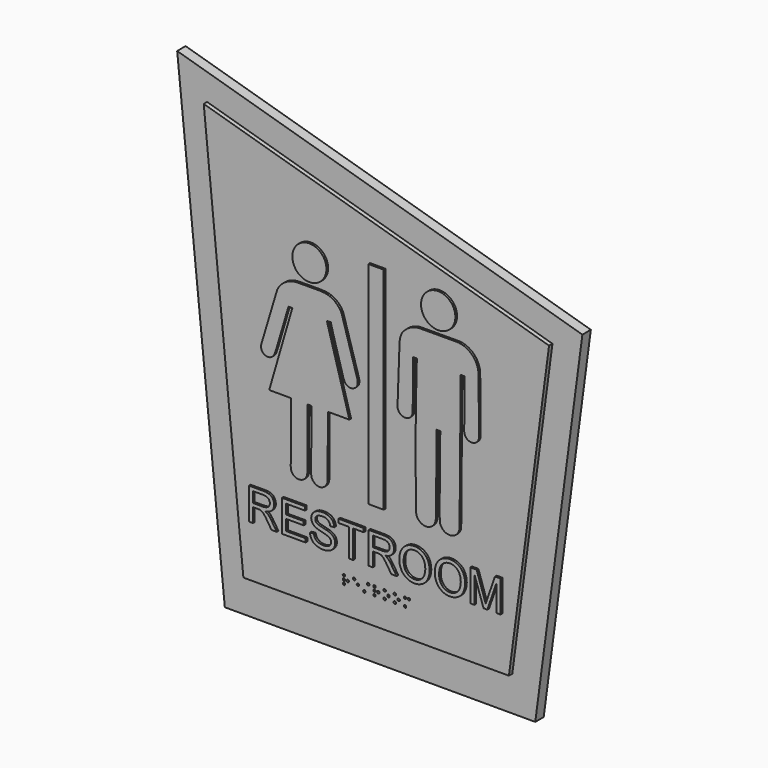
from build123d import *

# Parameters (mm, degrees)
F0_W     = 9.2540582
F0_H     = 127.1287526
F1_DEPTH = 6.35
F2_DEPTH = 8.89
F3_DEPTH = 10.16


with BuildPart() as f1:
    # F0 (on Front) → F1 (new body)
    with BuildSketch(Plane.XZ):
        Polygon((-261.8272132, -119.0471076), (-75.0463066, -119.023765), (-46.7040722, 95.3238632), (-290.4869222, 166.2895582), align=None)
        Polygon((-64.7140184, 84.666709), (-88.8685548, -98.010091), (-248.6300082, -97.9993468), (-272.4768744, 145.1469284), align=None, mode=Mode.SUBTRACT)
        Polygon((-248.6300082, -97.9993468), (-88.8685548, -98.010091), (-64.7140184, 84.666709), (-272.4768744, 145.1469284), align=None)
        Polygon((-231.562021, -85.1669112), (-232.4618668, -85.2533474), (-233.262297, -85.183345), (-234.0384194, -84.9753698), (-234.7665866, -84.6357464), (-235.2679064, -84.3007204), (-235.7212456, -83.9032104), (-236.296454, -83.205828), (-236.7232248, -82.4089284), (-236.9849464, -81.543652), (-237.0713318, -80.6438062), (-237.0013802, -79.843376), (-236.793405, -79.0672536), (-236.4537816, -78.3390864), (-236.1187556, -77.8377666), (-235.7212456, -77.3844274), (-235.0238632, -76.809219), (-234.2269636, -76.3824482), (-233.3617126, -76.1207266), (-232.4618414, -76.0343412), (-231.6614112, -76.1042928), (-230.8852888, -76.312268), (-230.1571216, -76.6518914), (-229.6558018, -76.9869174), (-229.2024626, -77.3844274), (-228.6272542, -78.0818098), (-228.2004834, -78.8787094), (-227.9387618, -79.7439604), (-227.8523764, -80.6438062), (-227.922328, -81.4442618), (-228.1303032, -82.2203842), (-228.4699266, -82.9485514), (-228.8049526, -83.4498712), (-229.2024626, -83.9032104), (-229.899845, -84.4783934), (-230.6967446, -84.9051896), align=None, mode=Mode.SUBTRACT)
        Polygon((-241.7956048, -66.4148024), (-244.3165548, -66.4148024), (-244.3165548, -47.3648024), (-235.8700896, -47.3648024), (-234.562269, -47.3849192), (-233.2656244, -47.5567756), (-231.9977072, -47.878111), (-231.3609038, -48.190658), (-230.7852128, -48.6051606), (-230.2867632, -49.1099348), (-229.8796012, -49.6908328), (-229.4376158, -50.5930408), (-229.1703062, -51.5614666), (-229.0869434, -52.562633), (-229.15499, -53.4977594), (-229.4038592, -54.40172), (-229.824026, -55.2398946), (-230.3993868, -55.980203), (-230.9028656, -56.4335422), (-231.4628848, -56.8148724), (-232.0691828, -57.1172086), (-233.2398942, -57.5138804), (-234.453684, -57.7474588), (-233.5732946, -58.2250042), (-232.9333162, -58.6960472), (-232.3759894, -59.2476336), (-231.8580326, -59.8363294), (-230.8411944, -61.230002), (-227.5275866, -66.4148024), (-230.6982686, -66.4148024), (-233.2191932, -62.451488), (-234.0998112, -61.1189278), (-235.0384428, -59.8265758), (-235.6278498, -59.1390232), (-236.3183996, -58.5531214), (-236.8722212, -58.2516234), (-237.46841, -58.0463406), (-238.033687, -57.9781162), (-238.8718362, -57.9553578), (-241.7956048, -57.9553578), align=None, mode=Mode.SUBTRACT)
        Polygon((-210.1445378, -66.4148024), (-224.3605876, -66.4148024), (-224.3605876, -47.3648024), (-210.5863708, -47.3648024), (-210.5863708, -49.6128802), (-221.8396376, -49.6128802), (-221.8396376, -55.4474126), (-211.301076, -55.4474126), (-211.301076, -57.6824856), (-221.8396376, -57.6824856), (-221.8396376, -64.16675), (-210.1445378, -64.16675), align=None, mode=Mode.SUBTRACT)
        Polygon((-207.519651, -60.294393), (-205.1416522, -60.0864686), (-205.0051526, -60.9067362), (-204.740891, -61.6951522), (-204.3554714, -62.4319808), (-203.8152642, -63.0453654), (-203.1685294, -63.545212), (-202.4387874, -63.9133596), (-201.7601248, -64.163321), (-201.0581196, -64.337311), (-200.2899474, -64.4448546), (-199.5150188, -64.4786366), (-198.6505044, -64.4412478), (-197.7971914, -64.2975854), (-196.9680846, -64.0498084), (-196.2710324, -63.7506218), (-195.6707034, -63.2869956), (-195.2049944, -62.6882414), (-194.9033948, -61.9922306), (-194.7850054, -61.2429814), (-194.8377104, -60.6860356), (-195.013961, -60.155074), (-195.304791, -59.6771476), (-195.6236626, -59.3408262), (-195.9934866, -59.0615278), (-196.4930792, -58.7796894), (-197.020053, -58.5531214), (-198.7036666, -58.0440546), (-200.4116388, -57.6240148), (-202.6434606, -57.0116462), (-203.3784096, -56.7537092), (-204.0891016, -56.4350154), (-204.7773654, -56.0434998), (-205.3908516, -55.5428912), (-205.9124406, -54.9471088), (-206.3275782, -54.2728404), (-206.6246566, -53.5388566), (-206.7514788, -52.9200872), (-206.7919664, -52.2897354), (-206.6989262, -51.3427472), (-206.422498, -50.4322334), (-205.973299, -49.593373), (-205.4925786, -48.9849922), (-204.9246854, -48.4570532), (-204.282929, -48.021875), (-203.5822954, -47.6896684), (-202.7649996, -47.4027246), (-201.922253, -47.2023948), (-201.0082594, -47.0789254), (-200.0867728, -47.0399618), (-198.8147408, -47.099982), (-197.5620128, -47.3287598), (-196.3508392, -47.722155), (-195.6218084, -48.0769676), (-194.954271, -48.5371648), (-194.36334, -49.0923072), (-193.8624012, -49.7298218), (-193.4781754, -50.412904), (-193.193162, -51.1429762), (-193.0074118, -51.9284458), (-192.9267922, -52.7315684), (-195.3437546, -52.9134832), (-195.4605692, -52.1453872), (-195.7272946, -51.4156706), (-196.1333898, -50.7533402), (-196.6627004, -50.1846342), (-197.3224146, -49.7655596), (-198.0547474, -49.492662), (-199.0110066, -49.3123474), (-199.9828106, -49.26203), (-200.9776016, -49.3065308), (-201.9596164, -49.4715546), (-202.6716038, -49.7128546), (-203.3159256, -50.1001538), (-203.756895, -50.5209302), (-204.1004554, -51.024409), (-204.2979404, -51.5566914), (-204.3619738, -52.1208254), (-204.3183112, -52.5982946), (-204.1768078, -53.0564344), (-203.9399274, -53.4633932), (-203.6212844, -53.8101032), (-202.9946918, -54.2051748), (-202.3072154, -54.4809426), (-201.0737914, -54.8606726), (-199.8203776, -55.168038), (-197.229603, -55.8193956), (-196.406897, -56.0731416), (-195.6036474, -56.3830216), (-194.670426, -56.8762642), (-193.8425384, -57.531127), (-193.147696, -58.3257152), (-192.8012654, -58.9352898), (-192.5531836, -59.591067), (-192.40246, -60.3059754), (-192.3550128, -61.0350824), (-192.4555206, -62.0411256), (-192.7494494, -63.0084846), (-193.2256486, -63.9003802), (-193.7307276, -64.5538968), (-194.324478, -65.1280638), (-194.9945808, -65.6109178), (-195.7271168, -65.992502), (-196.577585, -66.3224734), (-197.4602604, -66.5528768), (-198.4244698, -66.6950152), (-199.3980518, -66.7396684), (-200.8721662, -66.6843726), (-202.3255034, -66.4316172), (-203.731749, -65.9859996), (-204.5367258, -65.5792186), (-205.2725638, -65.057655), (-205.9229562, -64.4327896), (-206.4736028, -63.71844), (-206.9106352, -62.9391426), (-207.2321484, -62.1054892), (-207.4371772, -61.209682), align=None, mode=Mode.SUBTRACT)
        Polygon((-188.794263, -81.929859), (-188.8519718, -81.6433978), (-188.794263, -81.3569112), (-188.6325158, -81.1135538), (-188.389133, -80.9518066), (-188.1026718, -80.8940978), (-187.8162106, -80.9518066), (-187.5728532, -81.1135538), (-187.411106, -81.3569112), (-187.3533718, -81.6433978), (-187.411106, -81.929859), (-187.5728532, -82.1732164), (-187.8162106, -82.3349636), (-188.1026718, -82.3926978), (-188.389133, -82.3349636), (-188.6325158, -82.1732164), align=None, mode=Mode.SUBTRACT)
        Polygon((-188.794263, -79.643859), (-188.8519718, -79.3573978), (-188.794263, -79.0709112), (-188.6325158, -78.8275538), (-188.389133, -78.6658066), (-188.1026718, -78.6080978), (-187.8162106, -78.6658066), (-187.5728532, -78.8275538), (-187.411106, -79.0709112), (-187.3533718, -79.3573978), (-187.411106, -79.643859), (-187.5728532, -79.8872164), (-187.8162106, -80.0489636), (-188.1026718, -80.1066978), (-188.389133, -80.0489636), (-188.6325158, -79.8872164), align=None, mode=Mode.SUBTRACT)
        Polygon((-186.508263, -79.643859), (-186.5659718, -79.3573978), (-186.508263, -79.0709112), (-186.3465158, -78.8275538), (-186.103133, -78.6658066), (-185.8166718, -78.6080978), (-185.5302106, -78.6658066), (-185.2868532, -78.8275538), (-185.125106, -79.0709112), (-185.0673718, -79.3573978), (-185.125106, -79.643859), (-185.2868532, -79.8872164), (-185.5302106, -80.0489636), (-185.8166718, -80.1066978), (-186.103133, -80.0489636), (-186.3465158, -79.8872164), align=None, mode=Mode.SUBTRACT)
        Polygon((-188.816488, -77.357859), (-188.8742222, -77.0713978), (-188.816488, -76.7849112), (-188.6547408, -76.5415538), (-188.4113834, -76.3798066), (-188.1249222, -76.3220978), (-187.8384356, -76.3798066), (-187.5950782, -76.5415538), (-187.433331, -76.7849112), (-187.3756222, -77.0713978), (-187.433331, -77.357859), (-187.5950782, -77.6012164), (-187.8384356, -77.7629636), (-188.1249222, -77.8206978), (-188.4113834, -77.7629636), (-188.6547408, -77.6012164), align=None, mode=Mode.SUBTRACT)
        Polygon((-180.386863, -79.643859), (-180.4445718, -79.3573978), (-180.386863, -79.0709112), (-180.2251158, -78.8275538), (-179.981733, -78.6658066), (-179.6952718, -78.6080978), (-179.4088106, -78.6658066), (-179.1654532, -78.8275538), (-179.003706, -79.0709112), (-178.9459718, -79.3573978), (-179.003706, -79.643859), (-179.1654532, -79.8872164), (-179.4088106, -80.0489636), (-179.6952718, -80.1066978), (-179.981733, -80.0489636), (-180.2251158, -79.8872164), align=None, mode=Mode.SUBTRACT)
        Polygon((-182.695088, -77.357859), (-182.7528222, -77.0713978), (-182.695088, -76.7849112), (-182.5333408, -76.5415538), (-182.2899834, -76.3798066), (-182.0035222, -76.3220978), (-181.7170356, -76.3798066), (-181.4736782, -76.5415538), (-181.311931, -76.7849112), (-181.2542222, -77.0713978), (-181.311931, -77.357859), (-181.4736782, -77.6012164), (-181.7170356, -77.7629636), (-182.0035222, -77.8206978), (-182.2899834, -77.7629636), (-182.5333408, -77.6012164), align=None, mode=Mode.SUBTRACT)
        Polygon((-176.551463, -81.929859), (-176.6091718, -81.6433978), (-176.551463, -81.3569112), (-176.3897158, -81.1135538), (-176.146333, -80.9518066), (-175.8598718, -80.8940978), (-175.5734106, -80.9518066), (-175.3300532, -81.1135538), (-175.168306, -81.3569112), (-175.1105718, -81.6433978), (-175.168306, -81.929859), (-175.3300532, -82.1732164), (-175.5734106, -82.3349636), (-175.8598718, -82.3926978), (-176.146333, -82.3349636), (-176.3897158, -82.1732164), align=None, mode=Mode.SUBTRACT)
        Polygon((-170.430063, -81.929859), (-170.4877718, -81.6433978), (-170.430063, -81.3569112), (-170.2683158, -81.1135538), (-170.024933, -80.9518066), (-169.7384718, -80.8940978), (-169.4520106, -80.9518066), (-169.2086532, -81.1135538), (-169.046906, -81.3569112), (-168.9891718, -81.6433978), (-169.046906, -81.929859), (-169.2086532, -82.1732164), (-169.4520106, -82.3349636), (-169.7384718, -82.3926978), (-170.024933, -82.3349636), (-170.2683158, -82.1732164), align=None, mode=Mode.SUBTRACT)
        Polygon((-170.430063, -79.643859), (-170.4877718, -79.3573978), (-170.430063, -79.0709112), (-170.2683158, -78.8275538), (-170.024933, -78.6658066), (-169.7384718, -78.6080978), (-169.4520106, -78.6658066), (-169.2086532, -78.8275538), (-169.046906, -79.0709112), (-168.9891718, -79.3573978), (-169.046906, -79.643859), (-169.2086532, -79.8872164), (-169.4520106, -80.0489636), (-169.7384718, -80.1066978), (-170.024933, -80.0489636), (-170.2683158, -79.8872164), align=None, mode=Mode.SUBTRACT)
        Polygon((-174.243238, -77.380084), (-174.3009468, -77.0936228), (-174.243238, -76.8071616), (-174.0814908, -76.5637788), (-173.838108, -76.4020316), (-173.5516468, -76.3443228), (-173.2651856, -76.4020316), (-173.0218028, -76.5637788), (-172.8600556, -76.8071616), (-172.8023468, -77.0936228), (-172.8600556, -77.380084), (-173.0218028, -77.6234414), (-173.2651856, -77.785214), (-173.5516468, -77.8429228), (-173.838108, -77.785214), (-174.0814908, -77.6234414), align=None, mode=Mode.SUBTRACT)
        Polygon((-170.452288, -77.357859), (-170.5100222, -77.0713978), (-170.452288, -76.7849112), (-170.2905408, -76.5415538), (-170.0471834, -76.3798066), (-169.7607222, -76.3220978), (-169.4742356, -76.3798066), (-169.2308782, -76.5415538), (-169.069131, -76.7849112), (-169.0114222, -77.0713978), (-169.069131, -77.357859), (-169.2308782, -77.6012164), (-169.4742356, -77.7629636), (-169.7607222, -77.8206978), (-170.0471834, -77.7629636), (-170.2905408, -77.6012164), align=None, mode=Mode.SUBTRACT)
        Polygon((-181.5435536, -66.4148024), (-184.0645036, -66.4148024), (-184.0645036, -49.6128802), (-190.340869, -49.6128802), (-190.340869, -47.3648024), (-175.241204, -47.3648024), (-175.241204, -49.6128802), (-181.5435536, -49.6128802), align=None, mode=Mode.SUBTRACT)
        Polygon((-216.6317994, 69.5910216), (-215.6500386, 69.6736986), (-208.9904634, 69.7411356), (-203.294234, 69.7396116), (-202.2367304, 69.7333632), (-201.6876332, 69.7236858), (-201.4535214, 69.713602), (-200.5800662, 69.6334904), (-199.6147646, 69.6055504), (-198.6538826, 69.5090558), (-197.702297, 69.3444892), (-196.7648084, 69.1126634), (-195.846192, 68.8147976), (-194.951096, 68.4523396), (-194.0840162, 68.0271436), (-193.2493468, 67.541394), (-192.451355, 66.9975292), (-192.0808198, 66.638297), (-191.3264144, 65.9341582), (-190.9425188, 65.5892262), (-190.4337568, 65.0023592), (-189.9448576, 64.4016238), (-189.6397782, 63.9866132), (-189.2215926, 63.3366526), (-188.836554, 62.6636034), (-188.5884468, 62.208918), (-179.0511024, 30.3181512), (-178.9744706, 29.9642784), (-178.9094974, 29.6085768), (-178.863879, 29.2499034), (-178.8298938, 28.8894012), (-178.8476738, 28.5317946), (-178.8979404, 27.8175974), (-178.9304524, 27.4610068), (-179.1052298, 26.9211044), (-179.3508478, 26.4094976), (-179.662836, 25.9354574), (-180.0356064, 25.5075436), (-180.4623772, 25.1334778), (-180.9354522, 24.8200164), (-181.4462716, 24.5728236), (-181.985666, 24.3963698), (-182.543831, 24.29383), (-183.1106828, 24.2670838), (-183.676036, 24.3165884), (-184.229629, 24.4414802), (-184.7614796, 24.6394478), (-185.2619612, 24.9069606), (-185.7220822, 25.2391926), (-186.1334606, 25.6300986), (-186.4427818, 26.0376162), (-186.7149428, 26.4708386), (-186.94781, 26.9263876), (-187.13958, 27.4006818), (-187.2446598, 27.7264114), (-187.3555308, 28.0500582), (-187.4760792, 28.3702506), (-187.6024188, 28.6883348), (-188.4309668, 31.7338964), (-188.9034068, 33.371155), (-189.5917214, 35.7325422), (-191.8545312, 43.607101), (-193.1155396, 48.0314762), (-193.7319468, 50.2474738), (-194.3224968, 52.4704818), (-195.0269912, 55.2069762), (-195.6254406, 55.2170854), (-196.8224156, 55.2271438), (-197.4209412, 55.227093), (-183.8199524, 7.2196706), (-185.4896468, 7.2397874), (-188.3165144, 7.2470772), (-191.1434836, 7.2322944), (-196.7972188, 7.1995792), (-196.898133, -27.4675346), (-196.9182244, -29.3386764), (-196.9785494, -29.6607738), (-197.0683892, -30.2163988), (-197.211442, -30.7607716), (-197.406387, -31.2887868), (-197.65137, -31.7955168), (-197.944105, -32.2762626), (-198.2875384, -32.6724518), (-198.6683606, -33.032827), (-199.0828886, -33.353883), (-199.5270584, -33.6324702), (-199.9965774, -33.8658708), (-200.442703, -34.045398), (-200.9066086, -34.1720424), (-201.3820712, -34.2441784), (-201.8626646, -34.2607646), (-202.3419626, -34.2216486), (-202.8135136, -34.1272876), (-203.1395734, -34.0123018), (-203.463398, -33.891474), (-203.7834126, -33.7609434), (-204.1011412, -33.6245708), (-204.6090396, -33.3021686), (-205.0789396, -32.926528), (-205.5052532, -32.5020686), (-205.8829766, -32.033845), (-206.207614, -31.5273436), (-206.47533, -30.9886096), (-206.5696656, -30.6643024), (-206.6564828, -30.3388776), (-206.70647, -30.1207932), (-206.7588702, -29.8279312), (-206.7951414, -29.495115), (-206.8123626, -29.1595302), (-206.816579, -28.934791), (-206.8171886, -28.6345376), (-206.7773106, -15.2543764), (-206.7394138, -14.8023072), (-206.7166554, -14.3498824), (-206.7191192, -13.8968988), (-206.7367468, -13.4435596), (-206.6764218, 7.1392542), (-208.9299606, 7.1191374), (-209.0009536, -0.2647188), (-209.0304938, -7.6488544), (-209.0393076, -7.981188), (-209.0694574, -8.645271), (-209.0908188, -8.9770458), (-209.1109356, -28.7551876), (-209.1145932, -28.9630104), (-209.1282076, -29.169995), (-209.1554872, -29.3755826), (-209.1913774, -29.580332), (-209.2340494, -29.8954444), (-209.2875164, -30.2077374), (-209.3345064, -30.4129948), (-209.426429, -30.7153056), (-209.5363856, -31.0129428), (-209.6143636, -31.2101738), (-209.8093086, -31.6828932), (-210.0627244, -32.1270376), (-210.3704454, -32.5354188), (-210.7275186, -32.9014328), (-211.1281782, -33.2191614), (-211.5659218, -33.4834738), (-212.0490806, -33.7563206), (-212.5598746, -33.9731096), (-213.0918014, -34.1310722), (-213.63813, -34.2281764), (-214.207598, -34.2757252), (-214.7786408, -34.2544146), (-215.342978, -34.1645748), (-215.8924054, -34.0074758), (-216.4189474, -33.7854036), (-216.9149586, -33.5016094), (-217.3732, -33.160208), (-217.7870422, -32.7661524), (-218.1504654, -32.3251576), (-218.4582118, -31.8436498), (-218.7057856, -31.328614), (-218.88958, -30.7875432), (-218.9752796, -30.3388776), (-219.047949, -29.8890436), (-219.0827216, -29.5878758), (-219.1043878, -29.2475412), (-219.1117792, -28.9059366), (-219.1121602, -28.6777176), (-219.1111188, -28.3731208), (-219.0507938, 7.2196706), (-230.2599662, 7.2524874), (-230.9699978, 7.2574912), (-231.3581352, 7.2623172), (-231.500172, 7.2664066), (-231.618409, 7.274052), (-232.0280856, 7.3403206), (-231.9878774, 7.541768), (-218.145233, 55.227093), (-218.4068022, 55.204868), (-218.6683968, 55.1947588), (-218.929966, 55.204868), (-219.1915606, 55.227093), (-220.4792136, 55.227093), (-220.8616106, 53.8791404), (-221.3288182, 52.40401), (-221.779846, 50.9241044), (-222.203899, 49.436274), (-222.6117468, 47.943643), (-225.14306, 39.401369), (-227.347145, 31.9777364), (-227.6797072, 30.8739032), (-227.922201, 30.0853602), (-228.2644406, 29.036264), (-228.586284, 28.1340814), (-228.9296412, 27.2398236), (-229.1653786, 26.7570966), (-229.458266, 26.30678), (-229.8039092, 25.8955286), (-230.1971774, 25.5295654), (-230.64851, 25.188926), (-231.1425146, 24.9138186), (-231.6697678, 24.7095518), (-232.2201858, 24.5799864), (-232.7832022, 24.527637), (-233.3480474, 24.5534688), (-233.9039518, 24.6570246), (-234.440222, 24.8362978), (-234.9466218, 25.0878848), (-235.4134484, 25.4069342), (-235.8317864, 25.78735), (-236.1936094, 26.2218678), (-236.492034, 26.7021818), (-236.7212944, 27.2190718), (-236.8770218, 27.7626318), (-236.9403694, 28.4560772), (-236.9313524, 29.1523674), (-236.850047, 29.8439332), (-236.6973168, 30.5233324), (-236.4748636, 31.1831736), (-227.2997994, 61.8064042), (-226.8563408, 62.6862094), (-226.3500172, 63.5313944), (-225.783521, 64.3374888), (-225.1598494, 65.1002254), (-224.4823298, 65.8155402), (-223.7545182, 66.4796232), (-222.9803262, 67.0889946), (-222.1638178, 67.6404032), (-221.3093364, 68.1309026), (-220.421454, 68.557902), (-219.5048188, 68.9191662), (-218.5643076, 69.2127394), (-217.6049496, 69.4370976), align=None, mode=Mode.SUBTRACT)
        Polygon((-168.144063, -79.643859), (-168.2017718, -79.3573978), (-168.144063, -79.0709112), (-167.9823158, -78.8275538), (-167.738933, -78.6658066), (-167.4524718, -78.6080978), (-167.1660106, -78.6658066), (-166.9226532, -78.8275538), (-166.760906, -79.0709112), (-166.7031718, -79.3573978), (-166.760906, -79.643859), (-166.9226532, -79.8872164), (-167.1660106, -80.0489636), (-167.4524718, -80.1066978), (-167.738933, -80.0489636), (-167.9823158, -79.8872164), align=None, mode=Mode.SUBTRACT)
        Polygon((-164.308663, -81.929859), (-164.3663718, -81.6433978), (-164.308663, -81.3569112), (-164.1469158, -81.1135538), (-163.903533, -80.9518066), (-163.6170718, -80.8940978), (-163.3306106, -80.9518066), (-163.0872532, -81.1135538), (-162.925506, -81.3569112), (-162.8677718, -81.6433978), (-162.925506, -81.929859), (-163.0872532, -82.1732164), (-163.3306106, -82.3349636), (-163.6170718, -82.3926978), (-163.903533, -82.3349636), (-164.1469158, -82.1732164), align=None, mode=Mode.SUBTRACT)
        Polygon((-162.022663, -79.643859), (-162.0803718, -79.3573978), (-162.022663, -79.0709112), (-161.8609158, -78.8275538), (-161.617533, -78.6658066), (-161.3310718, -78.6080978), (-161.0446106, -78.6658066), (-160.8012532, -78.8275538), (-160.639506, -79.0709112), (-160.5817718, -79.3573978), (-160.639506, -79.643859), (-160.8012532, -79.8872164), (-161.0446106, -80.0489636), (-161.3310718, -80.1066978), (-161.617533, -80.0489636), (-161.8609158, -79.8872164), align=None, mode=Mode.SUBTRACT)
        Polygon((-164.330888, -77.357859), (-164.3886222, -77.0713978), (-164.330888, -76.7849112), (-164.1691408, -76.5415538), (-163.9257834, -76.3798066), (-163.6393222, -76.3220978), (-163.3528356, -76.3798066), (-163.1094782, -76.5415538), (-162.947731, -76.7849112), (-162.8900222, -77.0713978), (-162.947731, -77.357859), (-163.1094782, -77.6012164), (-163.3528356, -77.7629636), (-163.6393222, -77.8206978), (-163.9257834, -77.7629636), (-164.1691408, -77.6012164), align=None, mode=Mode.SUBTRACT)
        Polygon((-158.187263, -81.929859), (-158.2449718, -81.6433978), (-158.187263, -81.3569112), (-158.0255158, -81.1135538), (-157.782133, -80.9518066), (-157.4956718, -80.8940978), (-157.2092106, -80.9518066), (-156.9658532, -81.1135538), (-156.804106, -81.3569112), (-156.7463718, -81.6433978), (-156.804106, -81.929859), (-156.9658532, -82.1732164), (-157.2092106, -82.3349636), (-157.4956718, -82.3926978), (-157.782133, -82.3349636), (-158.0255158, -82.1732164), align=None, mode=Mode.SUBTRACT)
        Polygon((-155.901263, -79.643859), (-155.9589718, -79.3573978), (-155.901263, -79.0709112), (-155.7395158, -78.8275538), (-155.496133, -78.6658066), (-155.2096718, -78.6080978), (-154.9232106, -78.6658066), (-154.6798532, -78.8275538), (-154.518106, -79.0709112), (-154.4603718, -79.3573978), (-154.518106, -79.643859), (-154.6798532, -79.8872164), (-154.9232106, -80.0489636), (-155.2096718, -80.1066978), (-155.496133, -80.0489636), (-155.7395158, -79.8872164), align=None, mode=Mode.SUBTRACT)
        Polygon((-158.209488, -77.357859), (-158.2672222, -77.0713978), (-158.209488, -76.7849112), (-158.0477408, -76.5415538), (-157.8043834, -76.3798066), (-157.5179222, -76.3220978), (-157.2314356, -76.3798066), (-156.9880782, -76.5415538), (-156.826331, -76.7849112), (-156.7686222, -77.0713978), (-156.826331, -77.357859), (-156.9880782, -77.6012164), (-157.2314356, -77.7629636), (-157.5179222, -77.8206978), (-157.8043834, -77.7629636), (-158.0477408, -77.6012164), align=None, mode=Mode.SUBTRACT)
        Polygon((-152.065863, -81.929859), (-152.1235718, -81.6433978), (-152.065863, -81.3569112), (-151.9041158, -81.1135538), (-151.660733, -80.9518066), (-151.3742718, -80.8940978), (-151.0878106, -80.9518066), (-150.8444532, -81.1135538), (-150.682706, -81.3569112), (-150.6249718, -81.6433978), (-150.682706, -81.929859), (-150.8444532, -82.1732164), (-151.0878106, -82.3349636), (-151.3742718, -82.3926978), (-151.660733, -82.3349636), (-151.9041158, -82.1732164), align=None, mode=Mode.SUBTRACT)
        Polygon((-152.088088, -77.357859), (-152.1458222, -77.0713978), (-152.088088, -76.7849112), (-151.9263408, -76.5415538), (-151.6829834, -76.3798066), (-151.3965222, -76.3220978), (-151.1100356, -76.3798066), (-150.8666782, -76.5415538), (-150.704931, -76.7849112), (-150.6472222, -77.0713978), (-150.704931, -77.357859), (-150.8666782, -77.6012164), (-151.1100356, -77.7629636), (-151.3965222, -77.8206978), (-151.6829834, -77.7629636), (-151.9263408, -77.6012164), align=None, mode=Mode.SUBTRACT)
        Polygon((-149.757638, -77.380084), (-149.8153468, -77.0936228), (-149.757638, -76.8071616), (-149.5958908, -76.5637788), (-149.352508, -76.4020316), (-149.0660468, -76.3443228), (-148.7795856, -76.4020316), (-148.5362028, -76.5637788), (-148.3744556, -76.8071616), (-148.3167468, -77.0936228), (-148.3744556, -77.380084), (-148.5362028, -77.6234414), (-148.7795856, -77.785214), (-149.0660468, -77.8429228), (-149.352508, -77.785214), (-149.5958908, -77.6234414), align=None, mode=Mode.SUBTRACT)
        Polygon((-169.682795, -66.4148024), (-172.203745, -66.4148024), (-172.203745, -47.3648024), (-163.7572798, -47.3648024), (-162.4494592, -47.3849192), (-161.1528146, -47.5567756), (-159.8848974, -47.878111), (-159.248094, -48.190658), (-158.672403, -48.6051606), (-158.1739788, -49.1099348), (-157.7667914, -49.6908328), (-157.324806, -50.5930408), (-157.0574964, -51.5614666), (-156.9741336, -52.562633), (-157.0421802, -53.4977594), (-157.2910494, -54.40172), (-157.7112162, -55.2398946), (-158.286577, -55.980203), (-158.7900812, -56.4335422), (-159.350075, -56.8148724), (-159.956373, -57.1172086), (-161.1270844, -57.5138804), (-162.3408742, -57.7474588), (-161.4604848, -58.2250042), (-160.8205064, -58.6960472), (-160.2631796, -59.2476336), (-159.7452228, -59.8363294), (-158.7283846, -61.230002), (-155.4147768, -66.4148024), (-158.5854588, -66.4148024), (-161.1063834, -62.451488), (-161.9870014, -61.1189278), (-162.925633, -59.8265758), (-163.51504, -59.1390232), (-164.2055898, -58.5531214), (-164.7594114, -58.2516234), (-165.3556002, -58.0463406), (-165.9208772, -57.9781162), (-166.7590264, -57.9553578), (-169.682795, -57.9553578), align=None, mode=Mode.SUBTRACT)
        Polygon((-152.0326652, -50.6803406), (-151.243538, -49.71034), (-150.3706162, -48.9023406), (-149.3915478, -48.2269292), (-148.3262718, -47.6977964), (-147.139533, -47.315882), (-145.9133226, -47.0909904), (-144.6682908, -47.026957), (-143.4256212, -47.0944448), (-142.2037034, -47.3304616), (-141.0252704, -47.7306132), (-139.9122932, -48.287432), (-138.9188992, -48.9775246), (-138.0373668, -49.8057678), (-137.2867206, -50.7542292), (-136.6831404, -51.8024618), (-136.1928188, -52.9797264), (-135.849868, -54.2080704), (-135.638413, -55.554499), (-135.572119, -56.915812), (-135.6291928, -58.2553064), (-135.8455754, -59.5784432), (-136.2181426, -60.8663248), (-136.7416366, -62.1006378), (-137.3612188, -63.1467368), (-138.132439, -64.0866638), (-139.037441, -64.8985748), (-140.0552444, -65.5636738), (-141.1415008, -66.0754584), (-142.2837896, -66.4456888), (-143.4733478, -66.6676594), (-144.6812956, -66.7396684), (-145.9399926, -66.6717996), (-147.176871, -66.4288486), (-148.36775, -66.0156414), (-149.4892616, -65.4402298), (-150.4771438, -64.7382754), (-151.3532152, -63.9008882), (-152.09901, -62.9456958), (-152.6989326, -61.8927134), (-153.1749286, -60.758578), (-153.518235, -59.5775034), (-153.7243052, -58.3649074), (-153.7904722, -57.1367158), (-153.7341858, -55.706772), (-153.5210798, -54.2916872), (-153.1537196, -52.9086064), (-152.6738628, -51.753897), align=None, mode=Mode.SUBTRACT)
        Polygon((-130.6850066, -50.6803406), (-129.8958794, -49.71034), (-129.0229576, -48.9023406), (-128.0438892, -48.2269292), (-126.9786132, -47.6977964), (-125.7918744, -47.315882), (-124.565664, -47.0909904), (-123.3206322, -47.026957), (-122.0779626, -47.0944448), (-120.8560448, -47.3304616), (-119.6776118, -47.7306132), (-118.5646346, -48.287432), (-117.5712406, -48.9775246), (-116.6897082, -49.8057678), (-115.939062, -50.7542292), (-115.3354818, -51.8024618), (-114.8451602, -52.9797264), (-114.5022094, -54.2080704), (-114.2907544, -55.554499), (-114.2244604, -56.915812), (-114.2815342, -58.2553064), (-114.4979168, -59.5784432), (-114.870484, -60.8663248), (-115.393978, -62.1006378), (-116.0135602, -63.1467368), (-116.7847804, -64.0866638), (-117.6897824, -64.8985748), (-118.7075858, -65.5636738), (-119.7938422, -66.0754584), (-120.936131, -66.4456888), (-122.1256892, -66.6676594), (-123.333637, -66.7396684), (-124.592334, -66.6717996), (-125.8292124, -66.4288486), (-127.0200914, -66.0156414), (-128.141603, -65.4402298), (-129.1294852, -64.7382754), (-130.0055566, -63.9008882), (-130.7513514, -62.9456958), (-131.351274, -61.8927134), (-131.82727, -60.758578), (-132.1705764, -59.5775034), (-132.3766466, -58.3649074), (-132.4428136, -57.1367158), (-132.3865272, -55.706772), (-132.1734212, -54.2916872), (-131.8060864, -52.9086064), (-131.3262042, -51.753897), align=None, mode=Mode.SUBTRACT)
        Polygon((-104.1829514, -84.128483), (-105.0827972, -84.2149192), (-105.8832274, -84.1449168), (-106.6593498, -83.9369416), (-107.3875424, -83.5973436), (-107.8888368, -83.2623176), (-108.3422014, -82.8648076), (-108.9173844, -82.1674252), (-109.3441806, -81.3705256), (-109.6058768, -80.5052492), (-109.6922876, -79.6054034), (-109.6223106, -78.8049732), (-109.4143608, -78.0288508), (-109.0747374, -77.3006582), (-108.7397114, -76.7993638), (-108.3422014, -76.3459992), (-107.644819, -75.7708162), (-106.8479194, -75.34402), (-105.982643, -75.0823238), (-105.0827972, -74.995913), (-104.282367, -75.06589), (-103.5062446, -75.2738398), (-102.778052, -75.6134632), (-102.2767576, -75.9484892), (-101.823393, -76.3459992), (-101.24821, -77.0433816), (-100.8214138, -77.8402812), (-100.5597176, -78.7055576), (-100.4733068, -79.6054034), (-100.5432838, -80.4058336), (-100.7512336, -81.181956), (-101.090857, -81.9101486), (-101.425883, -82.411443), (-101.823393, -82.8648076), (-102.5208008, -83.4399906), (-103.317675, -83.8667614), align=None, mode=Mode.SUBTRACT)
        Polygon((-108.6238112, -66.4148024), (-111.0537784, -66.4148024), (-111.0537784, -47.3648024), (-107.259374, -47.3648024), (-102.7502898, -60.8531422), (-102.210997, -62.5002052), (-101.840665, -63.672974), (-101.4248416, -62.389766), (-100.827078, -60.619259), (-96.266, -47.3648024), (-92.8744142, -47.3648024), (-92.8744142, -66.4148024), (-95.3044068, -66.4148024), (-95.3044068, -50.4705112), (-100.8400828, -66.4148024), (-103.1141194, -66.4148024), (-108.6238112, -50.1976136), align=None, mode=Mode.SUBTRACT)
        Polygon((-142.0662386, 69.3641996), (-119.7830218, 69.4414664), (-118.7888404, 69.4359546), (-117.7978594, 69.3557668), (-116.815743, 69.2013348), (-115.8479776, 68.9735222), (-114.900075, 68.6736498), (-113.9773946, 68.3034194), (-113.085118, 67.864863), (-112.2283252, 67.3605206), (-111.4118676, 66.793237), (-110.6403426, 66.1661872), (-109.918119, 65.4829272), (-109.2492608, 64.7473432), (-108.637578, 63.9635754), (-108.086525, 63.1360688), (-107.5992006, 62.269497), (-107.1783734, 61.3687368), (-106.826431, 60.438919), (-106.5453546, 59.485276), (-106.336719, 58.5131926), (-106.255693, 57.9946008), (-106.1949108, 57.473215), (-106.155617, 56.9498988), (-106.13898, 56.4253634), (-105.8348912, 23.7521496), (-105.8405808, 23.1662986), (-105.92308, 22.5862642), (-106.0809664, 22.0220794), (-106.3114968, 21.4834724), (-106.6107088, 20.979765), (-106.9733954, 20.519644), (-107.3933082, 20.1111104), (-107.8631828, 19.7611746), (-108.3749166, 19.4759072), (-108.919645, 19.2602358), (-109.48797, 19.1178942), (-110.0700618, 19.0513462), (-110.6558366, 19.0617094), (-111.2351852, 19.1488568), (-111.7981, 19.311239), (-112.3348528, 19.5460874), (-112.8361472, 19.8492872), (-113.2933472, 20.2156568), (-113.698528, 20.6388208), (-114.0446792, 21.1115148), (-114.3258318, 21.6255092), (-114.5371344, 22.1719394), (-114.6749294, 22.741382), (-114.7229862, 23.0930704), (-114.740055, 23.4473496), (-114.6261106, 52.771294), (-116.8719024, 52.771294), (-117.5569912, -28.1019504), (-117.5670242, -28.7672526), (-117.651276, -29.4272716), (-117.8087052, -30.0737778), (-118.0373306, -30.6986432), (-118.334282, -31.2940954), (-118.6959018, -31.8526414), (-119.1175926, -32.3673216), (-119.5941474, -32.8316844), (-120.1195718, -33.2399386), (-120.6872872, -33.5869788), (-121.2901816, -33.8684616), (-121.920762, -34.0808564), (-122.571129, -34.2214962), (-123.2331038, -34.2886538), (-123.8984568, -34.2814656), (-124.5588314, -34.2000332), (-125.205998, -34.0453726), (-125.8318286, -33.8194142), (-126.4285254, -33.5249774), (-126.9886208, -33.1657706), (-127.505079, -32.7462642), (-127.9714992, -32.2716906), (-128.3819886, -31.7480442), (-128.7314418, -31.181802), (-129.01549, -30.5801014), (-129.2305772, -29.9504354), (-129.3739856, -29.300678), (-129.56413, -24.1437922), (-129.14503, 18.9952884), (-131.3146218, 19.013297), (-131.7905162, -28.1210004), (-131.9044606, -28.9581336), (-132.003419, -29.6189908), (-132.1763676, -30.2644302), (-132.4210458, -30.8862222), (-132.7343548, -31.4764166), (-133.1122814, -32.027495), (-133.550025, -32.5323708), (-134.0419468, -32.9845924), (-134.581773, -33.3784194), (-135.1625948, -33.7087718), (-135.7770208, -33.9714586), (-136.4171516, -34.1631016), (-137.0748338, -34.2812624), (-137.74166, -34.324417), (-138.4090704, -34.292032), (-139.0685814, -34.1844884), (-139.7117348, -34.0032086), (-140.330301, -33.7504786), (-140.9163806, -33.4295242), (-141.462506, -33.0444856), (-141.9616414, -32.6002396), (-142.4074622, -32.1025012), (-142.7942534, -31.557595), (-143.1170366, -30.9725314), (-143.3717224, -30.354778), (-143.5550596, -29.7121834), (-143.6646606, -29.053028), (-143.925036, -8.5761322), (-143.9863008, 11.899773), (-143.7156638, 32.3739764), (-143.2459162, 52.8471384), (-145.4342024, 52.8661884), (-145.7576968, 23.7521496), (-145.7956698, 23.155021), (-145.9114684, 22.5680016), (-146.1031368, 22.0011752), (-146.3673222, 21.4643208), (-146.6995542, 20.966684), (-147.0940416, 20.5168246), (-147.544028, 20.1224642), (-148.0417918, 19.79041), (-148.5787224, 19.526377), (-149.1455996, 19.3349118), (-149.7326698, 19.219291), (-150.3297984, 19.1815212), (-150.9267492, 19.2222628), (-151.5132352, 19.3407792), (-152.0791726, 19.5350638), (-152.6147824, 19.8017638), (-153.1108698, 20.1362564), (-153.5589004, 20.532852), (-153.951178, 20.9846672), (-154.2809208, 21.483955), (-154.5424646, 22.0221048), (-154.7313136, 22.5898456), (-154.8441912, 23.1774492), (-154.8792178, 23.7747556), (-153.6549886, 57.6812664), (-153.5925046, 58.6542896), (-153.4605262, 59.6203532), (-153.2584692, 60.5742248), (-152.9877814, 61.5109514), (-152.649936, 62.4256054), (-152.2466856, 63.3133608), (-151.6515382, 64.1425946), (-150.996015, 64.9249654), (-150.2837482, 65.656079), (-149.5187764, 66.3318206), (-148.7053668, 66.948431), (-147.8480914, 67.5024304), (-146.9517508, 67.9906946), (-146.0213742, 68.4105312), (-145.062194, 68.7595526), (-144.079595, 69.035803), (-143.0790636, 69.237733), align=None, mode=Mode.SUBTRACT)
        Polygon((-216.6724648, 77.2515854), (-216.9380218, 77.6814042), (-217.3116558, 78.4759162), (-217.618183, 79.2986476), (-217.8554952, 80.1439342), (-218.0219668, 81.0060102), (-218.1164294, 81.8788812), (-218.1382734, 82.7566036), (-218.0872956, 83.6330814), (-217.9639024, 84.5023456), (-217.8219672, 85.0524588), (-217.6651476, 85.5972126), (-217.5450056, 85.9547176), (-217.3353032, 86.4803198), (-217.100785, 86.9969558), (-216.9380218, 87.339043), (-216.6693406, 87.7619276), (-216.396316, 88.181942), (-216.1160016, 88.5971304), (-215.8313438, 89.0094486), (-215.2501156, 89.6508748), (-214.6172746, 90.2414248), (-213.937215, 90.776933), (-213.2147374, 91.253691), (-212.4549218, 91.6683206), (-211.6630768, 92.0179008), (-210.8447396, 92.3000186), (-210.005676, 92.5126928), (-209.1517534, 92.6543994), (-208.2889916, 92.7241478), (-207.423385, 92.7214808), (-206.561055, 92.6463984), (-205.7080468, 92.499434), (-204.870304, 92.2816036), (-204.0537194, 91.9944312), (-203.2640334, 91.6399742), (-202.5067832, 91.220671), (-201.7872774, 90.739468), (-201.6511588, 90.6066768), (-201.5129066, 90.476324), (-201.4184948, 90.391996), (-201.2726734, 90.2703808), (-201.123296, 90.1528296), (-201.0228136, 90.0755374), (-200.4129342, 89.4781802), (-199.855201, 88.8318772), (-199.3534748, 88.1412004), (-198.9113116, 87.4109504), (-198.5317848, 86.646258), (-198.2175614, 85.852508), (-197.9708766, 85.035263), (-197.7934068, 84.200238), (-197.686422, 83.353275), (-197.6506842, 82.500343), (-197.686422, 81.647411), (-197.7934068, 80.800448), (-197.9708766, 79.965423), (-198.2175614, 79.148178), (-198.5317848, 78.354428), (-198.9113116, 77.5897356), (-199.3534748, 76.8594856), (-199.855201, 76.1688088), (-200.4129342, 75.5225058), (-201.0228136, 74.9251486), (-201.1734102, 74.808969), (-201.3218732, 74.6903002), (-201.4185964, 74.6086138), (-201.5594394, 74.481182), (-201.696701, 74.3496354), (-201.7872774, 74.2608624), (-202.5113044, 73.7811834), (-203.272517, 73.3630486), (-204.065759, 73.0093536), (-204.8855186, 72.7225114), (-205.7262332, 72.5044778), (-206.5820862, 72.3567768), (-207.4472356, 72.2804244), (-208.3157124, 72.2759032), (-209.1816238, 72.3432894), (-210.0389754, 72.482075), (-210.8818744, 72.6913456), (-211.1151734, 72.7853764), (-211.3501488, 72.8747844), (-211.5878928, 72.9564708), (-211.8273386, 73.0335598), (-212.554312, 73.3786188), (-213.2535994, 73.7768654), (-213.9212892, 74.226039), (-214.5536984, 74.7236758), (-215.1473218, 75.2669818), (-215.3108978, 75.4550688), (-215.4785124, 75.6393458), (-215.6529088, 75.8171966), (-215.8313438, 75.9912374), (-216.1191512, 76.406502), (-216.4008626, 76.825729), align=None, mode=Mode.SUBTRACT)
        Polygon((-250.5700348, 115.3571226), (-251.4698806, 115.2706864), (-252.2703108, 115.3406888), (-253.0464332, 115.548664), (-253.7746258, 115.8882874), (-254.2759202, 116.2233134), (-254.7292848, 116.6208234), (-255.3044678, 117.3182058), (-255.731264, 118.1151054), (-255.9929602, 118.9803564), (-256.079371, 119.8802022), (-256.009394, 120.6806578), (-255.8014188, 121.4567802), (-255.4618208, 122.1849474), (-255.1267948, 122.6862672), (-254.7292848, 123.1396064), (-254.0319024, 123.7148148), (-253.2350028, 124.1415856), (-252.3697264, 124.4033072), (-251.4698806, 124.4896926), (-250.669425, 124.419741), (-249.893328, 124.2117658), (-249.1651354, 123.8721424), (-248.663841, 123.5371164), (-248.2104764, 123.1396064), (-247.6352934, 122.442224), (-247.2084972, 121.6453244), (-246.946801, 120.7800734), (-246.8603902, 119.8802022), (-246.9303672, 119.079772), (-247.138317, 118.3036496), (-247.4779404, 117.5754824), (-247.8129664, 117.0741626), (-248.2104764, 116.6208234), (-248.9078588, 116.0456404), (-249.7047584, 115.6188442), align=None, mode=Mode.SUBTRACT)
        with Locations((-167.8070177, 29.8195365)):
            Rectangle(F0_W, F0_H, mode=Mode.SUBTRACT)
        Polygon((-140.691108, 81.5700934), (-140.7190734, 82.3711078), (-140.6838182, 83.191477), (-140.5845296, 84.0065884), (-140.419455, 84.815934), (-140.1899406, 85.60943), (-139.868021, 86.4510844), (-139.4738892, 87.261446), (-139.0105678, 88.0343172), (-138.4815874, 88.7638306), (-137.8909866, 89.4443982), (-137.2432358, 90.0708638), (-136.5433388, 90.6384268), (-135.7965788, 91.1427692), (-135.0086454, 91.5800302), (-134.1856092, 91.9468824), (-133.3336678, 92.2405318), (-132.4593744, 92.4587432), (-131.5693838, 92.5998402), (-130.6704524, 92.662756), (-129.769489, 92.647008), (-128.8733262, 92.5527232), (-127.9887966, 92.3806128), (-127.1226566, 92.1319976), (-126.2815102, 91.8087572), (-125.4717836, 91.4133554), (-124.6996236, 90.9488402), (-123.9709484, 90.4187168), (-123.3459306, 89.8786112), (-122.7661248, 89.2902456), (-122.2352394, 88.6573792), (-121.7567034, 87.9840506), (-121.3335648, 87.2746032), (-120.9685668, 86.5335836), (-120.6639954, 85.7657416), (-120.4218318, 84.9759794), (-120.2448192, 84.1741522), (-120.1310018, 83.3609458), (-120.0820052, 82.5609474), (-120.0956704, 81.7595266), (-120.1806334, 80.8947328), (-120.3380118, 80.0401244), (-120.5667642, 79.2017974), (-120.8652142, 78.3856954), (-121.2312536, 77.5975842), (-121.6622916, 76.8430518), (-122.1553056, 76.127483), (-122.7067396, 75.455907), (-123.3127328, 74.833099), (-123.9689672, 74.2634532), (-124.6707692, 73.751059), (-125.440821, 73.2843848), (-126.2486426, 72.8866208), (-127.0880364, 72.5607896), (-127.952627, 72.3093296), (-128.8358612, 72.134222), (-129.731008, 72.0367622), (-130.6312348, 72.0177122), (-131.5296836, 72.0771736), (-132.4195472, 72.21474), (-133.2940184, 72.42937), (-134.1464424, 72.7193872), (-134.9703676, 73.0826072), (-135.7594948, 73.5162614), (-136.5078042, 74.0170478), (-137.2096062, 74.5811564), (-137.8595922, 75.2042946), (-138.4527584, 75.8817126), (-138.9846344, 76.6082796), (-139.4511562, 77.378433), (-139.8487678, 78.1863054), (-140.1744212, 79.0257754), (-140.4257034, 79.8904168), (-140.6006332, 80.7737018), align=None, mode=Mode.SUBTRACT)
        Polygon((-84.3014824, 66.8496504), (-85.2013282, 66.7632142), (-86.0017838, 66.8332166), (-86.7778808, 67.0411918), (-87.5060734, 67.3808152), (-88.0073932, 67.7158412), (-88.4607324, 68.1133512), (-89.0359408, 68.8107336), (-89.4627116, 69.6076332), (-89.7244332, 70.4728842), (-89.8108186, 71.3727554), (-89.7408416, 72.1731856), (-89.5328918, 72.949308), (-89.1932684, 73.6774752), (-88.8582424, 74.178795), (-88.4607324, 74.6321342), (-87.76335, 75.2073426), (-86.9664504, 75.6341134), (-86.101174, 75.895835), (-85.2013282, 75.9822204), (-84.400898, 75.9122688), (-83.6247756, 75.7042936), (-82.896583, 75.3646702), (-82.3952886, 75.0296442), (-81.9419494, 74.6321342), (-81.366741, 73.9347518), (-80.9399702, 73.1378522), (-80.6782486, 72.2726012), (-80.5918378, 71.3727554), (-80.6618148, 70.5722998), (-80.86979, 69.7961774), (-81.2094134, 69.0680102), (-81.5444394, 68.5666904), (-81.941924, 68.1133512), (-82.6393318, 67.5381682), (-83.4362314, 67.111372), align=None, mode=Mode.SUBTRACT)
        Polygon((-208.9904634, 69.7411356), (-215.6500386, 69.6736986), (-216.6317994, 69.5910216), (-217.6049496, 69.4370976), (-218.5643076, 69.2127394), (-219.5048188, 68.9191662), (-220.421454, 68.557902), (-221.3093364, 68.1309026), (-222.1638178, 67.6404032), (-222.9803262, 67.0889946), (-223.7545182, 66.4796232), (-224.4823298, 65.8155402), (-225.1598494, 65.1002254), (-225.783521, 64.3374888), (-226.3500172, 63.5313944), (-226.8563408, 62.6862094), (-227.2997994, 61.8064042), (-236.4748636, 31.1831736), (-236.6973168, 30.5233324), (-236.850047, 29.8439332), (-236.9313524, 29.1523674), (-236.9403694, 28.4560772), (-236.8770218, 27.7626318), (-236.7212944, 27.2190718), (-236.492034, 26.7021818), (-236.1936094, 26.2218678), (-235.8317864, 25.78735), (-235.4134484, 25.4069342), (-234.9466218, 25.0878848), (-234.440222, 24.8362978), (-233.9039518, 24.6570246), (-233.3480474, 24.5534688), (-232.7832022, 24.527637), (-232.2201858, 24.5799864), (-231.6697678, 24.7095518), (-231.1425146, 24.9138186), (-230.64851, 25.188926), (-230.1971774, 25.5295654), (-229.8039092, 25.8955286), (-229.458266, 26.30678), (-229.1653786, 26.7570966), (-228.9296412, 27.2398236), (-228.586284, 28.1340814), (-228.2644406, 29.036264), (-227.922201, 30.0853602), (-227.6797072, 30.8739032), (-227.347145, 31.9777364), (-225.14306, 39.401369), (-222.6117468, 47.943643), (-222.203899, 49.436274), (-221.779846, 50.9241044), (-221.3288182, 52.40401), (-220.8616106, 53.8791404), (-220.4792136, 55.227093), (-219.1915606, 55.227093), (-218.929966, 55.204868), (-218.6683968, 55.1947588), (-218.4068022, 55.204868), (-218.145233, 55.227093), (-231.9878774, 7.541768), (-232.0280856, 7.3403206), (-231.618409, 7.274052), (-231.500172, 7.2664066), (-231.3581352, 7.2623172), (-230.9699978, 7.2574912), (-230.2599662, 7.2524874), (-219.0507938, 7.2196706), (-219.1111188, -28.3731208), (-219.1121602, -28.6777176), (-219.1117792, -28.9059366), (-219.1043878, -29.2475412), (-219.0827216, -29.5878758), (-219.047949, -29.8890436), (-218.9752796, -30.3388776), (-218.88958, -30.7875432), (-218.7057856, -31.328614), (-218.4582118, -31.8436498), (-218.1504654, -32.3251576), (-217.7870422, -32.7661524), (-217.3732, -33.160208), (-216.9149586, -33.5016094), (-216.4189474, -33.7854036), (-215.8924054, -34.0074758), (-215.342978, -34.1645748), (-214.7786408, -34.2544146), (-214.207598, -34.2757252), (-213.63813, -34.2281764), (-213.0918014, -34.1310722), (-212.5598746, -33.9731096), (-212.0490806, -33.7563206), (-211.5659218, -33.4834738), (-211.1281782, -33.2191614), (-210.7275186, -32.9014328), (-210.3704454, -32.5354188), (-210.0627244, -32.1270376), (-209.8093086, -31.6828932), (-209.6143636, -31.2101738), (-209.5363856, -31.0129428), (-209.426429, -30.7153056), (-209.3345064, -30.4129948), (-209.2875164, -30.2077374), (-209.2340494, -29.8954444), (-209.1913774, -29.580332), (-209.1554872, -29.3755826), (-209.1282076, -29.169995), (-209.1145932, -28.9630104), (-209.1109356, -28.7551876), (-209.0908188, -8.9770458), (-209.0694574, -8.645271), (-209.0393076, -7.981188), (-209.0304938, -7.6488544), (-209.0009536, -0.2647188), (-208.9299606, 7.1191374), (-206.6764218, 7.1392542), (-206.7367468, -13.4435596), (-206.7191192, -13.8968988), (-206.7166554, -14.3498824), (-206.7394138, -14.8023072), (-206.7773106, -15.2543764), (-206.8171886, -28.6345376), (-206.816579, -28.934791), (-206.8123626, -29.1595302), (-206.7951414, -29.495115), (-206.7588702, -29.8279312), (-206.70647, -30.1207932), (-206.6564828, -30.3388776), (-206.5696656, -30.6643024), (-206.47533, -30.9886096), (-206.207614, -31.5273436), (-205.8829766, -32.033845), (-205.5052532, -32.5020686), (-205.0789396, -32.926528), (-204.6090396, -33.3021686), (-204.1011412, -33.6245708), (-203.7834126, -33.7609434), (-203.463398, -33.891474), (-203.1395734, -34.0123018), (-202.8135136, -34.1272876), (-202.3419626, -34.2216486), (-201.8626646, -34.2607646), (-201.3820712, -34.2441784), (-200.9066086, -34.1720424), (-200.442703, -34.045398), (-199.9965774, -33.8658708), (-199.5270584, -33.6324702), (-199.0828886, -33.353883), (-198.6683606, -33.032827), (-198.2875384, -32.6724518), (-197.944105, -32.2762626), (-197.65137, -31.7955168), (-197.406387, -31.2887868), (-197.211442, -30.7607716), (-197.0683892, -30.2163988), (-196.9785494, -29.6607738), (-196.9182244, -29.3386764), (-196.898133, -27.4675346), (-196.7972188, 7.1995792), (-191.1434836, 7.2322944), (-188.3165144, 7.2470772), (-185.4896468, 7.2397874), (-183.8199524, 7.2196706), (-197.4209412, 55.227093), (-196.8224156, 55.2271438), (-195.6254406, 55.2170854), (-195.0269912, 55.2069762), (-194.3224968, 52.4704818), (-193.7319468, 50.2474738), (-193.1155396, 48.0314762), (-191.8545312, 43.607101), (-189.5917214, 35.7325422), (-188.9034068, 33.371155), (-188.4309668, 31.7338964), (-187.6024188, 28.6883348), (-187.4760792, 28.3702506), (-187.3555308, 28.0500582), (-187.2446598, 27.7264114), (-187.13958, 27.4006818), (-186.94781, 26.9263876), (-186.7149428, 26.4708386), (-186.4427818, 26.0376162), (-186.1334606, 25.6300986), (-185.7220822, 25.2391926), (-185.2619612, 24.9069606), (-184.7614796, 24.6394478), (-184.229629, 24.4414802), (-183.676036, 24.3165884), (-183.1106828, 24.2670838), (-182.543831, 24.29383), (-181.985666, 24.3963698), (-181.4462716, 24.5728236), (-180.9354522, 24.8200164), (-180.4623772, 25.1334778), (-180.0356064, 25.5075436), (-179.662836, 25.9354574), (-179.3508478, 26.4094976), (-179.1052298, 26.9211044), (-178.9304524, 27.4610068), (-178.8979404, 27.8175974), (-178.8476738, 28.5317946), (-178.8298938, 28.8894012), (-178.863879, 29.2499034), (-178.9094974, 29.6085768), (-178.9744706, 29.9642784), (-179.0511024, 30.3181512), (-188.5884468, 62.208918), (-188.836554, 62.6636034), (-189.2215926, 63.3366526), (-189.6397782, 63.9866132), (-189.9448576, 64.4016238), (-190.4337568, 65.0023592), (-190.9425188, 65.5892262), (-191.3264144, 65.9341582), (-192.0808198, 66.638297), (-192.451355, 66.9975292), (-193.2493468, 67.541394), (-194.0840162, 68.0271436), (-194.951096, 68.4523396), (-195.846192, 68.8147976), (-196.7648084, 69.1126634), (-197.702297, 69.3444892), (-198.6538826, 69.5090558), (-199.6147646, 69.6055504), (-200.5800662, 69.6334904), (-201.4535214, 69.713602), (-201.6876332, 69.7236858), (-202.2367304, 69.7333632), (-203.294234, 69.7396116), align=None)
        Polygon((-118.7888404, 69.4359546), (-119.7830218, 69.4414664), (-142.0662386, 69.3641996), (-143.0790636, 69.237733), (-144.079595, 69.035803), (-145.062194, 68.7595526), (-146.0213742, 68.4105312), (-146.9517508, 67.9906946), (-147.8480914, 67.5024304), (-148.7053668, 66.948431), (-149.5187764, 66.3318206), (-150.2837482, 65.656079), (-150.996015, 64.9249654), (-151.6515382, 64.1425946), (-152.2466856, 63.3133608), (-152.649936, 62.4256054), (-152.9877814, 61.5109514), (-153.2584692, 60.5742248), (-153.4605262, 59.6203532), (-153.5925046, 58.6542896), (-153.6549886, 57.6812664), (-154.8792178, 23.7747556), (-154.8441912, 23.1774492), (-154.7313136, 22.5898456), (-154.5424646, 22.0221048), (-154.2809208, 21.483955), (-153.951178, 20.9846672), (-153.5589004, 20.532852), (-153.1108698, 20.1362564), (-152.6147824, 19.8017638), (-152.0791726, 19.5350638), (-151.5132352, 19.3407792), (-150.9267492, 19.2222628), (-150.3297984, 19.1815212), (-149.7326698, 19.219291), (-149.1455996, 19.3349118), (-148.5787224, 19.526377), (-148.0417918, 19.79041), (-147.544028, 20.1224642), (-147.0940416, 20.5168246), (-146.6995542, 20.966684), (-146.3673222, 21.4643208), (-146.1031368, 22.0011752), (-145.9114684, 22.5680016), (-145.7956698, 23.155021), (-145.7576968, 23.7521496), (-145.4342024, 52.8661884), (-143.2459162, 52.8471384), (-143.7156638, 32.3739764), (-143.9863008, 11.899773), (-143.925036, -8.5761322), (-143.6646606, -29.053028), (-143.5550596, -29.7121834), (-143.3717224, -30.354778), (-143.1170366, -30.9725314), (-142.7942534, -31.557595), (-142.4074622, -32.1025012), (-141.9616414, -32.6002396), (-141.462506, -33.0444856), (-140.9163806, -33.4295242), (-140.330301, -33.7504786), (-139.7117348, -34.0032086), (-139.0685814, -34.1844884), (-138.4090704, -34.292032), (-137.74166, -34.324417), (-137.0748338, -34.2812624), (-136.4171516, -34.1631016), (-135.7770208, -33.9714586), (-135.1625948, -33.7087718), (-134.581773, -33.3784194), (-134.0419468, -32.9845924), (-133.550025, -32.5323708), (-133.1122814, -32.027495), (-132.7343548, -31.4764166), (-132.4210458, -30.8862222), (-132.1763676, -30.2644302), (-132.003419, -29.6189908), (-131.9044606, -28.9581336), (-131.7905162, -28.1210004), (-131.3146218, 19.013297), (-129.14503, 18.9952884), (-129.56413, -24.1437922), (-129.3739856, -29.300678), (-129.2305772, -29.9504354), (-129.01549, -30.5801014), (-128.7314418, -31.181802), (-128.3819886, -31.7480442), (-127.9714992, -32.2716906), (-127.505079, -32.7462642), (-126.9886208, -33.1657706), (-126.4285254, -33.5249774), (-125.8318286, -33.8194142), (-125.205998, -34.0453726), (-124.5588314, -34.2000332), (-123.8984568, -34.2814656), (-123.2331038, -34.2886538), (-122.571129, -34.2214962), (-121.920762, -34.0808564), (-121.2901816, -33.8684616), (-120.6872872, -33.5869788), (-120.1195718, -33.2399386), (-119.5941474, -32.8316844), (-119.1175926, -32.3673216), (-118.6959018, -31.8526414), (-118.334282, -31.2940954), (-118.0373306, -30.6986432), (-117.8087052, -30.0737778), (-117.651276, -29.4272716), (-117.5670242, -28.7672526), (-117.5569912, -28.1019504), (-116.8719024, 52.771294), (-114.6261106, 52.771294), (-114.740055, 23.4473496), (-114.7229862, 23.0930704), (-114.6749294, 22.741382), (-114.5371344, 22.1719394), (-114.3258318, 21.6255092), (-114.0446792, 21.1115148), (-113.698528, 20.6388208), (-113.2933472, 20.2156568), (-112.8361472, 19.8492872), (-112.3348528, 19.5460874), (-111.7981, 19.311239), (-111.2351852, 19.1488568), (-110.6558366, 19.0617094), (-110.0700618, 19.0513462), (-109.48797, 19.1178942), (-108.919645, 19.2602358), (-108.3749166, 19.4759072), (-107.8631828, 19.7611746), (-107.3933082, 20.1111104), (-106.9733954, 20.519644), (-106.6107088, 20.979765), (-106.3114968, 21.4834724), (-106.0809664, 22.0220794), (-105.92308, 22.5862642), (-105.8405808, 23.1662986), (-105.8348912, 23.7521496), (-106.13898, 56.4253634), (-106.155617, 56.9498988), (-106.1949108, 57.473215), (-106.255693, 57.9946008), (-106.336719, 58.5131926), (-106.5453546, 59.485276), (-106.826431, 60.438919), (-107.1783734, 61.3687368), (-107.5992006, 62.269497), (-108.086525, 63.1360688), (-108.637578, 63.9635754), (-109.2492608, 64.7473432), (-109.918119, 65.4829272), (-110.6403426, 66.1661872), (-111.4118676, 66.793237), (-112.2283252, 67.3605206), (-113.085118, 67.864863), (-113.9773946, 68.3034194), (-114.900075, 68.6736498), (-115.8479776, 68.9735222), (-116.815743, 69.2013348), (-117.7978594, 69.3557668), align=None)
        with Locations((-167.8070177, 29.8195365)):
            Rectangle(F0_W, F0_H)
        Polygon((-140.6838182, 83.191477), (-140.7190734, 82.3711078), (-140.691108, 81.5700934), (-140.6006332, 80.7737018), (-140.4257034, 79.8904168), (-140.1744212, 79.0257754), (-139.8487678, 78.1863054), (-139.4511562, 77.378433), (-138.9846344, 76.6082796), (-138.4527584, 75.8817126), (-137.8595922, 75.2042946), (-137.2096062, 74.5811564), (-136.5078042, 74.0170478), (-135.7594948, 73.5162614), (-134.9703676, 73.0826072), (-134.1464424, 72.7193872), (-133.2940184, 72.42937), (-132.4195472, 72.21474), (-131.5296836, 72.0771736), (-130.6312348, 72.0177122), (-129.731008, 72.0367622), (-128.8358612, 72.134222), (-127.952627, 72.3093296), (-127.0880364, 72.5607896), (-126.2486426, 72.8866208), (-125.440821, 73.2843848), (-124.6707692, 73.751059), (-123.9689672, 74.2634532), (-123.3127328, 74.833099), (-122.7067396, 75.455907), (-122.1553056, 76.127483), (-121.6622916, 76.8430518), (-121.2312536, 77.5975842), (-120.8652142, 78.3856954), (-120.5667642, 79.2017974), (-120.3380118, 80.0401244), (-120.1806334, 80.8947328), (-120.0956704, 81.7595266), (-120.0820052, 82.5609474), (-120.1310018, 83.3609458), (-120.2448192, 84.1741522), (-120.4218318, 84.9759794), (-120.6639954, 85.7657416), (-120.9685668, 86.5335836), (-121.3335648, 87.2746032), (-121.7567034, 87.9840506), (-122.2352394, 88.6573792), (-122.7661248, 89.2902456), (-123.3459306, 89.8786112), (-123.9709484, 90.4187168), (-124.6996236, 90.9488402), (-125.4717836, 91.4133554), (-126.2815102, 91.8087572), (-127.1226566, 92.1319976), (-127.9887966, 92.3806128), (-128.8733262, 92.5527232), (-129.769489, 92.647008), (-130.6704524, 92.662756), (-131.5693838, 92.5998402), (-132.4593744, 92.4587432), (-133.3336678, 92.2405318), (-134.1856092, 91.9468824), (-135.0086454, 91.5800302), (-135.7965788, 91.1427692), (-136.5433388, 90.6384268), (-137.2432358, 90.0708638), (-137.8909866, 89.4443982), (-138.4815874, 88.7638306), (-139.0105678, 88.0343172), (-139.4738892, 87.261446), (-139.868021, 86.4510844), (-140.1899406, 85.60943), (-140.419455, 84.815934), (-140.5845296, 84.0065884), align=None)
        Polygon((-217.3116558, 78.4759162), (-216.9380218, 77.6814042), (-216.6724648, 77.2515854), (-216.4008626, 76.825729), (-216.1191512, 76.406502), (-215.8313438, 75.9912374), (-215.6529088, 75.8171966), (-215.4785124, 75.6393458), (-215.3108978, 75.4550688), (-215.1473218, 75.2669818), (-214.5536984, 74.7236758), (-213.9212892, 74.226039), (-213.2535994, 73.7768654), (-212.554312, 73.3786188), (-211.8273386, 73.0335598), (-211.5878928, 72.9564708), (-211.3501488, 72.8747844), (-211.1151734, 72.7853764), (-210.8818744, 72.6913456), (-210.0389754, 72.482075), (-209.1816238, 72.3432894), (-208.3157124, 72.2759032), (-207.4472356, 72.2804244), (-206.5820862, 72.3567768), (-205.7262332, 72.5044778), (-204.8855186, 72.7225114), (-204.065759, 73.0093536), (-203.272517, 73.3630486), (-202.5113044, 73.7811834), (-201.7872774, 74.2608624), (-201.696701, 74.3496354), (-201.5594394, 74.481182), (-201.4185964, 74.6086138), (-201.3218732, 74.6903002), (-201.1734102, 74.808969), (-201.0228136, 74.9251486), (-200.4129342, 75.5225058), (-199.855201, 76.1688088), (-199.3534748, 76.8594856), (-198.9113116, 77.5897356), (-198.5317848, 78.354428), (-198.2175614, 79.148178), (-197.9708766, 79.965423), (-197.7934068, 80.800448), (-197.686422, 81.647411), (-197.6506842, 82.500343), (-197.686422, 83.353275), (-197.7934068, 84.200238), (-197.9708766, 85.035263), (-198.2175614, 85.852508), (-198.5317848, 86.646258), (-198.9113116, 87.4109504), (-199.3534748, 88.1412004), (-199.855201, 88.8318772), (-200.4129342, 89.4781802), (-201.0228136, 90.0755374), (-201.123296, 90.1528296), (-201.2726734, 90.2703808), (-201.4184948, 90.391996), (-201.5129066, 90.476324), (-201.6511588, 90.6066768), (-201.7872774, 90.739468), (-202.5067832, 91.220671), (-203.2640334, 91.6399742), (-204.0537194, 91.9944312), (-204.870304, 92.2816036), (-205.7080468, 92.499434), (-206.561055, 92.6463984), (-207.423385, 92.7214808), (-208.2889916, 92.7241478), (-209.1517534, 92.6543994), (-210.005676, 92.5126928), (-210.8447396, 92.3000186), (-211.6630768, 92.0179008), (-212.4549218, 91.6683206), (-213.2147374, 91.253691), (-213.937215, 90.776933), (-214.6172746, 90.2414248), (-215.2501156, 89.6508748), (-215.8313438, 89.0094486), (-216.1160016, 88.5971304), (-216.396316, 88.181942), (-216.6693406, 87.7619276), (-216.9380218, 87.339043), (-217.100785, 86.9969558), (-217.3353032, 86.4803198), (-217.5450056, 85.9547176), (-217.6651476, 85.5972126), (-217.8219672, 85.0524588), (-217.9639024, 84.5023456), (-218.0872956, 83.6330814), (-218.1382734, 82.7566036), (-218.1164294, 81.8788812), (-218.0219668, 81.0060102), (-217.8554952, 80.1439342), (-217.618183, 79.2986476), align=None)
        Polygon((-129.0229576, -48.9023406), (-129.8958794, -49.71034), (-130.6850066, -50.6803406), (-131.3262042, -51.753897), (-131.8060864, -52.9086064), (-132.1734212, -54.2916872), (-132.3865272, -55.706772), (-132.4428136, -57.1367158), (-132.3766466, -58.3649074), (-132.1705764, -59.5775034), (-131.82727, -60.758578), (-131.351274, -61.8927134), (-130.7513514, -62.9456958), (-130.0055566, -63.9008882), (-129.1294852, -64.7382754), (-128.141603, -65.4402298), (-127.0200914, -66.0156414), (-125.8292124, -66.4288486), (-124.592334, -66.6717996), (-123.333637, -66.7396684), (-122.1256892, -66.6676594), (-120.936131, -66.4456888), (-119.7938422, -66.0754584), (-118.7075858, -65.5636738), (-117.6897824, -64.8985748), (-116.7847804, -64.0866638), (-116.0135602, -63.1467368), (-115.393978, -62.1006378), (-114.870484, -60.8663248), (-114.4979168, -59.5784432), (-114.2815342, -58.2553064), (-114.2244604, -56.915812), (-114.2907544, -55.554499), (-114.5022094, -54.2080704), (-114.8451602, -52.9797264), (-115.3354818, -51.8024618), (-115.939062, -50.7542292), (-116.6897082, -49.8057678), (-117.5712406, -48.9775246), (-118.5646346, -48.287432), (-119.6776118, -47.7306132), (-120.8560448, -47.3304616), (-122.0779626, -47.0944448), (-123.3206322, -47.026957), (-124.565664, -47.0909904), (-125.7918744, -47.315882), (-126.9786132, -47.6977964), (-128.0438892, -48.2269292), align=None)
        Polygon((-127.3683254, -63.1924822), (-127.9921748, -62.6009162), (-128.5653004, -61.8873286), (-129.031365, -61.0996238), (-129.3809706, -60.2537784), (-129.6477214, -59.24677), (-129.8026614, -58.2166222), (-129.8438856, -57.1757048), (-129.8070048, -55.9330606), (-129.645664, -54.7003986), (-129.3614634, -53.490114), (-129.0210526, -52.593621), (-128.5339568, -51.7675622), (-127.9141968, -51.0357628), (-127.1334008, -50.383821), (-126.2597678, -49.8627908), (-125.3150656, -49.4857024), (-124.3227638, -49.2619284), (-123.3076528, -49.1970568), (-122.403616, -49.2547402), (-121.516013, -49.4358168), (-120.6867538, -49.7355876), (-119.9095646, -50.1521476), (-119.1901858, -50.6881892), (-118.5581322, -51.3248402), (-118.0273484, -52.0481052), (-117.6095438, -52.8420076), (-117.1550108, -54.1535874), (-116.891181, -55.5163736), (-116.823363, -56.9028072), (-116.862987, -58.0029574), (-117.0167586, -59.0930238), (-117.2830522, -60.1611954), (-117.6239202, -61.031882), (-118.0868352, -61.8442756), (-118.6620944, -62.5814344), (-119.4306984, -63.2966476), (-120.3108846, -63.8690366), (-121.2764148, -64.2814818), (-122.29846, -64.521715), (-123.3466164, -64.5825734), (-124.219208, -64.5338816), (-125.07722, -64.3677148), (-125.9049298, -64.0871718), (-126.668022, -63.6911604), align=None, mode=Mode.SUBTRACT)
        Polygon((-150.3706162, -48.9023406), (-151.243538, -49.71034), (-152.0326652, -50.6803406), (-152.6738628, -51.753897), (-153.1537196, -52.9086064), (-153.5210798, -54.2916872), (-153.7341858, -55.706772), (-153.7904722, -57.1367158), (-153.7243052, -58.3649074), (-153.518235, -59.5775034), (-153.1749286, -60.758578), (-152.6989326, -61.8927134), (-152.09901, -62.9456958), (-151.3532152, -63.9008882), (-150.4771438, -64.7382754), (-149.4892616, -65.4402298), (-148.36775, -66.0156414), (-147.176871, -66.4288486), (-145.9399926, -66.6717996), (-144.6812956, -66.7396684), (-143.4733478, -66.6676594), (-142.2837896, -66.4456888), (-141.1415008, -66.0754584), (-140.0552444, -65.5636738), (-139.037441, -64.8985748), (-138.132439, -64.0866638), (-137.3612188, -63.1467368), (-136.7416366, -62.1006378), (-136.2181426, -60.8663248), (-135.8455754, -59.5784432), (-135.6291928, -58.2553064), (-135.572119, -56.915812), (-135.638413, -55.554499), (-135.849868, -54.2080704), (-136.1928188, -52.9797264), (-136.6831404, -51.8024618), (-137.2867206, -50.7542292), (-138.0373668, -49.8057678), (-138.9188992, -48.9775246), (-139.9122932, -48.287432), (-141.0252704, -47.7306132), (-142.2037034, -47.3304616), (-143.4256212, -47.0944448), (-144.6682908, -47.026957), (-145.9133226, -47.0909904), (-147.139533, -47.315882), (-148.3262718, -47.6977964), (-149.3915478, -48.2269292), align=None)
        Polygon((-148.715984, -63.1924822), (-149.3398334, -62.6009162), (-149.912959, -61.8873286), (-150.3790236, -61.0996238), (-150.7286292, -60.2537784), (-150.99538, -59.24677), (-151.15032, -58.2166222), (-151.1915442, -57.1757048), (-151.1546634, -55.9330606), (-150.9933226, -54.7003986), (-150.709122, -53.490114), (-150.3687112, -52.593621), (-149.8816154, -51.7675622), (-149.2618554, -51.0357628), (-148.4810594, -50.383821), (-147.6074264, -49.8627908), (-146.6627242, -49.4857024), (-145.6704224, -49.2619284), (-144.6553114, -49.1970568), (-143.7512746, -49.2547402), (-142.8636716, -49.4358168), (-142.0344124, -49.7355876), (-141.2572232, -50.1521476), (-140.5378444, -50.6881892), (-139.9057908, -51.3248402), (-139.375007, -52.0481052), (-138.9572024, -52.8420076), (-138.5026694, -54.1535874), (-138.2388396, -55.5163736), (-138.1710216, -56.9028072), (-138.2106456, -58.0029574), (-138.3644172, -59.0930238), (-138.6307108, -60.1611954), (-138.9715788, -61.031882), (-139.4344938, -61.8442756), (-140.009753, -62.5814344), (-140.778357, -63.2966476), (-141.6585432, -63.8690366), (-142.6240734, -64.2814818), (-143.6461186, -64.521715), (-144.694275, -64.5825734), (-145.5668666, -64.5338816), (-146.4248786, -64.3677148), (-147.2525884, -64.0871718), (-148.0156806, -63.6911604), align=None, mode=Mode.SUBTRACT)
        Polygon((-244.3165548, -47.3648024), (-244.3165548, -66.4148024), (-241.7956048, -66.4148024), (-241.7956048, -57.9553578), (-238.8718362, -57.9553578), (-238.033687, -57.9781162), (-237.46841, -58.0463406), (-236.8722212, -58.2516234), (-236.3183996, -58.5531214), (-235.6278498, -59.1390232), (-235.0384428, -59.8265758), (-234.0998112, -61.1189278), (-233.2191932, -62.451488), (-230.6982686, -66.4148024), (-227.5275866, -66.4148024), (-230.8411944, -61.230002), (-231.8580326, -59.8363294), (-232.3759894, -59.2476336), (-232.9333162, -58.6960472), (-233.5732946, -58.2250042), (-234.453684, -57.7474588), (-233.2398942, -57.5138804), (-232.0691828, -57.1172086), (-231.4628848, -56.8148724), (-230.9028656, -56.4335422), (-230.3993868, -55.980203), (-229.824026, -55.2398946), (-229.4038592, -54.40172), (-229.15499, -53.4977594), (-229.0869434, -52.562633), (-229.1703062, -51.5614666), (-229.4376158, -50.5930408), (-229.8796012, -49.6908328), (-230.2867632, -49.1099348), (-230.7852128, -48.6051606), (-231.3609038, -48.190658), (-231.9977072, -47.878111), (-233.2656244, -47.5567756), (-234.562269, -47.3849192), (-235.8700896, -47.3648024), align=None)
        Polygon((-236.3768704, -55.7722786), (-241.7956048, -55.7722786), (-241.7956048, -49.469929), (-235.7661274, -49.469929), (-234.8418214, -49.5164872), (-233.9322728, -49.6875816), (-233.2623732, -49.9419372), (-232.6669464, -50.3405648), (-232.2412932, -50.799873), (-231.9266888, -51.3413502), (-231.7385002, -51.9386312), (-231.685846, -52.562633), (-231.741853, -53.1617428), (-231.9129474, -53.7386276), (-232.1926268, -54.271418), (-232.5974774, -54.7594282), (-233.0993814, -55.1468798), (-233.6740056, -55.414926), (-234.5596528, -55.6352456), (-235.4644008, -55.7548542), align=None, mode=Mode.SUBTRACT)
        Polygon((-172.203745, -47.3648024), (-172.203745, -66.4148024), (-169.682795, -66.4148024), (-169.682795, -57.9553578), (-166.7590264, -57.9553578), (-165.9208772, -57.9781162), (-165.3556002, -58.0463406), (-164.7594114, -58.2516234), (-164.2055898, -58.5531214), (-163.51504, -59.1390232), (-162.925633, -59.8265758), (-161.9870014, -61.1189278), (-161.1063834, -62.451488), (-158.5854588, -66.4148024), (-155.4147768, -66.4148024), (-158.7283846, -61.230002), (-159.7452228, -59.8363294), (-160.2631796, -59.2476336), (-160.8205064, -58.6960472), (-161.4604848, -58.2250042), (-162.3408742, -57.7474588), (-161.1270844, -57.5138804), (-159.956373, -57.1172086), (-159.350075, -56.8148724), (-158.7900812, -56.4335422), (-158.286577, -55.980203), (-157.7112162, -55.2398946), (-157.2910494, -54.40172), (-157.0421802, -53.4977594), (-156.9741336, -52.562633), (-157.0574964, -51.5614666), (-157.324806, -50.5930408), (-157.7667914, -49.6908328), (-158.1739788, -49.1099348), (-158.672403, -48.6051606), (-159.248094, -48.190658), (-159.8848974, -47.878111), (-161.1528146, -47.5567756), (-162.4494592, -47.3849192), (-163.7572798, -47.3648024), align=None)
        Polygon((-164.2640606, -55.7722786), (-169.682795, -55.7722786), (-169.682795, -49.469929), (-163.6533176, -49.469929), (-162.7290116, -49.5164872), (-161.819463, -49.6875816), (-161.1495634, -49.9419372), (-160.5541366, -50.3405648), (-160.1284834, -50.799873), (-159.8139044, -51.3413502), (-159.6256904, -51.9386312), (-159.5730362, -52.562633), (-159.6290432, -53.1617428), (-159.8001376, -53.7386276), (-160.079817, -54.271418), (-160.4846676, -54.7594282), (-160.986597, -55.1468798), (-161.5611958, -55.414926), (-162.446843, -55.6352456), (-163.3516164, -55.7548542), align=None, mode=Mode.SUBTRACT)
        Polygon((-111.0537784, -47.3648024), (-111.0537784, -66.4148024), (-108.6238112, -66.4148024), (-108.6238112, -50.1976136), (-103.1141194, -66.4148024), (-100.8400828, -66.4148024), (-95.3044068, -50.4705112), (-95.3044068, -66.4148024), (-92.8744142, -66.4148024), (-92.8744142, -47.3648024), (-96.266, -47.3648024), (-100.827078, -60.619259), (-101.4248416, -62.389766), (-101.840665, -63.672974), (-102.210997, -62.5002052), (-102.7502898, -60.8531422), (-107.259374, -47.3648024), align=None)
        Polygon((-128.5653004, -61.8873286), (-127.9921748, -62.6009162), (-127.3683254, -63.1924822), (-126.668022, -63.6911604), (-125.9049298, -64.0871718), (-125.07722, -64.3677148), (-124.219208, -64.5338816), (-123.3466164, -64.5825734), (-122.29846, -64.521715), (-121.2764148, -64.2814818), (-120.3108846, -63.8690366), (-119.4306984, -63.2966476), (-118.6620944, -62.5814344), (-118.0868352, -61.8442756), (-117.6239202, -61.031882), (-117.2830522, -60.1611954), (-117.0167586, -59.0930238), (-116.862987, -58.0029574), (-116.823363, -56.9028072), (-116.891181, -55.5163736), (-117.1550108, -54.1535874), (-117.6095438, -52.8420076), (-118.0273484, -52.0481052), (-118.5581322, -51.3248402), (-119.1901858, -50.6881892), (-119.9095646, -50.1521476), (-120.6867538, -49.7355876), (-121.516013, -49.4358168), (-122.403616, -49.2547402), (-123.3076528, -49.1970568), (-124.3227638, -49.2619284), (-125.3150656, -49.4857024), (-126.2597678, -49.8627908), (-127.1334008, -50.383821), (-127.9141968, -51.0357628), (-128.5339568, -51.7675622), (-129.0210526, -52.593621), (-129.3614634, -53.490114), (-129.645664, -54.7003986), (-129.8070048, -55.9330606), (-129.8438856, -57.1757048), (-129.8026614, -58.2166222), (-129.6477214, -59.24677), (-129.3809706, -60.2537784), (-129.031365, -61.0996238), align=None)
        Polygon((-149.912959, -61.8873286), (-149.3398334, -62.6009162), (-148.715984, -63.1924822), (-148.0156806, -63.6911604), (-147.2525884, -64.0871718), (-146.4248786, -64.3677148), (-145.5668666, -64.5338816), (-144.694275, -64.5825734), (-143.6461186, -64.521715), (-142.6240734, -64.2814818), (-141.6585432, -63.8690366), (-140.778357, -63.2966476), (-140.009753, -62.5814344), (-139.4344938, -61.8442756), (-138.9715788, -61.031882), (-138.6307108, -60.1611954), (-138.3644172, -59.0930238), (-138.2106456, -58.0029574), (-138.1710216, -56.9028072), (-138.2388396, -55.5163736), (-138.5026694, -54.1535874), (-138.9572024, -52.8420076), (-139.375007, -52.0481052), (-139.9057908, -51.3248402), (-140.5378444, -50.6881892), (-141.2572232, -50.1521476), (-142.0344124, -49.7355876), (-142.8636716, -49.4358168), (-143.7512746, -49.2547402), (-144.6553114, -49.1970568), (-145.6704224, -49.2619284), (-146.6627242, -49.4857024), (-147.6074264, -49.8627908), (-148.4810594, -50.383821), (-149.2618554, -51.0357628), (-149.8816154, -51.7675622), (-150.3687112, -52.593621), (-150.709122, -53.490114), (-150.9933226, -54.7003986), (-151.1546634, -55.9330606), (-151.1915442, -57.1757048), (-151.15032, -58.2166222), (-150.99538, -59.24677), (-150.7286292, -60.2537784), (-150.3790236, -61.0996238), align=None)
        Polygon((-224.3605876, -47.3648024), (-224.3605876, -66.4148024), (-210.1445378, -66.4148024), (-210.1445378, -64.16675), (-221.8396376, -64.16675), (-221.8396376, -57.6824856), (-211.301076, -57.6824856), (-211.301076, -55.4474126), (-221.8396376, -55.4474126), (-221.8396376, -49.6128802), (-210.5863708, -49.6128802), (-210.5863708, -47.3648024), align=None)
        Polygon((-205.0051526, -60.9067362), (-205.1416522, -60.0864686), (-207.519651, -60.294393), (-207.4371772, -61.209682), (-207.2321484, -62.1054892), (-206.9106352, -62.9391426), (-206.4736028, -63.71844), (-205.9229562, -64.4327896), (-205.2725638, -65.057655), (-204.5367258, -65.5792186), (-203.731749, -65.9859996), (-202.3255034, -66.4316172), (-200.8721662, -66.6843726), (-199.3980518, -66.7396684), (-198.4244698, -66.6950152), (-197.4602604, -66.5528768), (-196.577585, -66.3224734), (-195.7271168, -65.992502), (-194.9945808, -65.6109178), (-194.324478, -65.1280638), (-193.7307276, -64.5538968), (-193.2256486, -63.9003802), (-192.7494494, -63.0084846), (-192.4555206, -62.0411256), (-192.3550128, -61.0350824), (-192.40246, -60.3059754), (-192.5531836, -59.591067), (-192.8012654, -58.9352898), (-193.147696, -58.3257152), (-193.8425384, -57.531127), (-194.670426, -56.8762642), (-195.6036474, -56.3830216), (-196.406897, -56.0731416), (-197.229603, -55.8193956), (-199.8203776, -55.168038), (-201.0737914, -54.8606726), (-202.3072154, -54.4809426), (-202.9946918, -54.2051748), (-203.6212844, -53.8101032), (-203.9399274, -53.4633932), (-204.1768078, -53.0564344), (-204.3183112, -52.5982946), (-204.3619738, -52.1208254), (-204.2979404, -51.5566914), (-204.1004554, -51.024409), (-203.756895, -50.5209302), (-203.3159256, -50.1001538), (-202.6716038, -49.7128546), (-201.9596164, -49.4715546), (-200.9776016, -49.3065308), (-199.9828106, -49.26203), (-199.0110066, -49.3123474), (-198.0547474, -49.492662), (-197.3224146, -49.7655596), (-196.6627004, -50.1846342), (-196.1333898, -50.7533402), (-195.7272946, -51.4156706), (-195.4605692, -52.1453872), (-195.3437546, -52.9134832), (-192.9267922, -52.7315684), (-193.0074118, -51.9284458), (-193.193162, -51.1429762), (-193.4781754, -50.412904), (-193.8624012, -49.7298218), (-194.36334, -49.0923072), (-194.954271, -48.5371648), (-195.6218084, -48.0769676), (-196.3508392, -47.722155), (-197.5620128, -47.3287598), (-198.8147408, -47.099982), (-200.0867728, -47.0399618), (-201.0082594, -47.0789254), (-201.922253, -47.2023948), (-202.7649996, -47.4027246), (-203.5822954, -47.6896684), (-204.282929, -48.021875), (-204.9246854, -48.4570532), (-205.4925786, -48.9849922), (-205.973299, -49.593373), (-206.422498, -50.4322334), (-206.6989262, -51.3427472), (-206.7919664, -52.2897354), (-206.7514788, -52.9200872), (-206.6246566, -53.5388566), (-206.3275782, -54.2728404), (-205.9124406, -54.9471088), (-205.3908516, -55.5428912), (-204.7773654, -56.0434998), (-204.0891016, -56.4350154), (-203.3784096, -56.7537092), (-202.6434606, -57.0116462), (-200.4116388, -57.6240148), (-198.7036666, -58.0440546), (-197.020053, -58.5531214), (-196.4930792, -58.7796894), (-195.9934866, -59.0615278), (-195.6236626, -59.3408262), (-195.304791, -59.6771476), (-195.013961, -60.155074), (-194.8377104, -60.6860356), (-194.7850054, -61.2429814), (-194.9033948, -61.9922306), (-195.2049944, -62.6882414), (-195.6707034, -63.2869956), (-196.2710324, -63.7506218), (-196.9680846, -64.0498084), (-197.7971914, -64.2975854), (-198.6505044, -64.4412478), (-199.5150188, -64.4786366), (-200.2899474, -64.4448546), (-201.0581196, -64.337311), (-201.7601248, -64.163321), (-202.4387874, -63.9133596), (-203.1685294, -63.545212), (-203.8152642, -63.0453654), (-204.3554714, -62.4319808), (-204.740891, -61.6951522), align=None)
        Polygon((-184.0645036, -49.6128802), (-184.0645036, -66.4148024), (-181.5435536, -66.4148024), (-181.5435536, -49.6128802), (-175.241204, -49.6128802), (-175.241204, -47.3648024), (-190.340869, -47.3648024), (-190.340869, -49.6128802), align=None)
        Polygon((-105.8832274, -84.1449168), (-105.0827972, -84.2149192), (-104.1829514, -84.128483), (-103.317675, -83.8667614), (-102.5208008, -83.4399906), (-101.823393, -82.8648076), (-101.425883, -82.411443), (-101.090857, -81.9101486), (-100.7512336, -81.181956), (-100.5432838, -80.4058336), (-100.4733068, -79.6054034), (-100.5597176, -78.7055576), (-100.8214138, -77.8402812), (-101.24821, -77.0433816), (-101.823393, -76.3459992), (-102.2767576, -75.9484892), (-102.778052, -75.6134632), (-103.5062446, -75.2738398), (-104.282367, -75.06589), (-105.0827972, -74.995913), (-105.982643, -75.0823238), (-106.8479194, -75.34402), (-107.644819, -75.7708162), (-108.3422014, -76.3459992), (-108.7397114, -76.7993638), (-109.0747374, -77.3006582), (-109.4143608, -78.0288508), (-109.6223106, -78.8049732), (-109.6922876, -79.6054034), (-109.6058768, -80.5052492), (-109.3441806, -81.3705256), (-108.9173844, -82.1674252), (-108.3422014, -82.8648076), (-107.8888368, -83.2623176), (-107.3875424, -83.5973436), (-106.6593498, -83.9369416), align=None)
        Polygon((-252.2703108, 115.3406888), (-251.4698806, 115.2706864), (-250.5700348, 115.3571226), (-249.7047584, 115.6188442), (-248.9078588, 116.0456404), (-248.2104764, 116.6208234), (-247.8129664, 117.0741626), (-247.4779404, 117.5754824), (-247.138317, 118.3036496), (-246.9303672, 119.079772), (-246.8603902, 119.8802022), (-246.946801, 120.7800734), (-247.2084972, 121.6453244), (-247.6352934, 122.442224), (-248.2104764, 123.1396064), (-248.663841, 123.5371164), (-249.1651354, 123.8721424), (-249.893328, 124.2117658), (-250.669425, 124.419741), (-251.4698806, 124.4896926), (-252.3697264, 124.4033072), (-253.2350028, 124.1415856), (-254.0319024, 123.7148148), (-254.7292848, 123.1396064), (-255.1267948, 122.6862672), (-255.4618208, 122.1849474), (-255.8014188, 121.4567802), (-256.009394, 120.6806578), (-256.079371, 119.8802022), (-255.9929602, 118.9803564), (-255.731264, 118.1151054), (-255.3044678, 117.3182058), (-254.7292848, 116.6208234), (-254.2759202, 116.2233134), (-253.7746258, 115.8882874), (-253.0464332, 115.548664), align=None)
        Polygon((-86.0017838, 66.8332166), (-85.2013282, 66.7632142), (-84.3014824, 66.8496504), (-83.4362314, 67.111372), (-82.6393318, 67.5381682), (-81.941924, 68.1133512), (-81.5444394, 68.5666904), (-81.2094134, 69.0680102), (-80.86979, 69.7961774), (-80.6618148, 70.5722998), (-80.5918378, 71.3727554), (-80.6782486, 72.2726012), (-80.9399702, 73.1378522), (-81.366741, 73.9347518), (-81.9419494, 74.6321342), (-82.3952886, 75.0296442), (-82.896583, 75.3646702), (-83.6247756, 75.7042936), (-84.400898, 75.9122688), (-85.2013282, 75.9822204), (-86.101174, 75.895835), (-86.9664504, 75.6341134), (-87.76335, 75.2073426), (-88.4607324, 74.6321342), (-88.8582424, 74.178795), (-89.1932684, 73.6774752), (-89.5328918, 72.949308), (-89.7408416, 72.1731856), (-89.8108186, 71.3727554), (-89.7244332, 70.4728842), (-89.4627116, 69.6076332), (-89.0359408, 68.8107336), (-88.4607324, 68.1133512), (-88.0073932, 67.7158412), (-87.5060734, 67.3808152), (-86.7778808, 67.0411918), align=None)
        Polygon((-233.262297, -85.183345), (-232.4618668, -85.2533474), (-231.562021, -85.1669112), (-230.6967446, -84.9051896), (-229.899845, -84.4783934), (-229.2024626, -83.9032104), (-228.8049526, -83.4498712), (-228.4699266, -82.9485514), (-228.1303032, -82.2203842), (-227.922328, -81.4442618), (-227.8523764, -80.6438062), (-227.9387618, -79.7439604), (-228.2004834, -78.8787094), (-228.6272542, -78.0818098), (-229.2024626, -77.3844274), (-229.6558018, -76.9869174), (-230.1571216, -76.6518914), (-230.8852888, -76.312268), (-231.6614112, -76.1042928), (-232.4618414, -76.0343412), (-233.3617126, -76.1207266), (-234.2269636, -76.3824482), (-235.0238632, -76.809219), (-235.7212456, -77.3844274), (-236.1187556, -77.8377666), (-236.4537816, -78.3390864), (-236.793405, -79.0672536), (-237.0013802, -79.843376), (-237.0713318, -80.6438062), (-236.9849464, -81.543652), (-236.7232248, -82.4089284), (-236.296454, -83.205828), (-235.7212456, -83.9032104), (-235.2679064, -84.3007204), (-234.7665866, -84.6357464), (-234.0384194, -84.9753698), align=None)
        Polygon((-241.7956048, -49.469929), (-241.7956048, -55.7722786), (-236.3768704, -55.7722786), (-235.4644008, -55.7548542), (-234.5596528, -55.6352456), (-233.6740056, -55.414926), (-233.0993814, -55.1468798), (-232.5974774, -54.7594282), (-232.1926268, -54.271418), (-231.9129474, -53.7386276), (-231.741853, -53.1617428), (-231.685846, -52.562633), (-231.7385002, -51.9386312), (-231.9266888, -51.3413502), (-232.2412932, -50.799873), (-232.6669464, -50.3405648), (-233.2623732, -49.9419372), (-233.9322728, -49.6875816), (-234.8418214, -49.5164872), (-235.7661274, -49.469929), align=None)
        Polygon((-169.682795, -49.469929), (-169.682795, -55.7722786), (-164.2640606, -55.7722786), (-163.3516164, -55.7548542), (-162.446843, -55.6352456), (-161.5611958, -55.414926), (-160.986597, -55.1468798), (-160.4846676, -54.7594282), (-160.079817, -54.271418), (-159.8001376, -53.7386276), (-159.6290432, -53.1617428), (-159.5730362, -52.562633), (-159.6256904, -51.9386312), (-159.8139044, -51.3413502), (-160.1284834, -50.799873), (-160.5541366, -50.3405648), (-161.1495634, -49.9419372), (-161.819463, -49.6875816), (-162.7290116, -49.5164872), (-163.6533176, -49.469929), align=None)
        Polygon((-174.243238, -76.8071616), (-174.3009468, -77.0936228), (-174.243238, -77.380084), (-174.0814908, -77.6234414), (-173.838108, -77.785214), (-173.5516468, -77.8429228), (-173.2651856, -77.785214), (-173.0218028, -77.6234414), (-172.8600556, -77.380084), (-172.8023468, -77.0936228), (-172.8600556, -76.8071616), (-173.0218028, -76.5637788), (-173.2651856, -76.4020316), (-173.5516468, -76.3443228), (-173.838108, -76.4020316), (-174.0814908, -76.5637788), align=None)
        Polygon((-149.757638, -76.8071616), (-149.8153468, -77.0936228), (-149.757638, -77.380084), (-149.5958908, -77.6234414), (-149.352508, -77.785214), (-149.0660468, -77.8429228), (-148.7795856, -77.785214), (-148.5362028, -77.6234414), (-148.3744556, -77.380084), (-148.3167468, -77.0936228), (-148.3744556, -76.8071616), (-148.5362028, -76.5637788), (-148.7795856, -76.4020316), (-149.0660468, -76.3443228), (-149.352508, -76.4020316), (-149.5958908, -76.5637788), align=None)
        Polygon((-158.209488, -76.7849112), (-158.2672222, -77.0713978), (-158.209488, -77.357859), (-158.0477408, -77.6012164), (-157.8043834, -77.7629636), (-157.5179222, -77.8206978), (-157.2314356, -77.7629636), (-156.9880782, -77.6012164), (-156.826331, -77.357859), (-156.7686222, -77.0713978), (-156.826331, -76.7849112), (-156.9880782, -76.5415538), (-157.2314356, -76.3798066), (-157.5179222, -76.3220978), (-157.8043834, -76.3798066), (-158.0477408, -76.5415538), align=None)
        Polygon((-188.816488, -76.7849112), (-188.8742222, -77.0713978), (-188.816488, -77.357859), (-188.6547408, -77.6012164), (-188.4113834, -77.7629636), (-188.1249222, -77.8206978), (-187.8384356, -77.7629636), (-187.5950782, -77.6012164), (-187.433331, -77.357859), (-187.3756222, -77.0713978), (-187.433331, -76.7849112), (-187.5950782, -76.5415538), (-187.8384356, -76.3798066), (-188.1249222, -76.3220978), (-188.4113834, -76.3798066), (-188.6547408, -76.5415538), align=None)
        Polygon((-152.088088, -76.7849112), (-152.1458222, -77.0713978), (-152.088088, -77.357859), (-151.9263408, -77.6012164), (-151.6829834, -77.7629636), (-151.3965222, -77.8206978), (-151.1100356, -77.7629636), (-150.8666782, -77.6012164), (-150.704931, -77.357859), (-150.6472222, -77.0713978), (-150.704931, -76.7849112), (-150.8666782, -76.5415538), (-151.1100356, -76.3798066), (-151.3965222, -76.3220978), (-151.6829834, -76.3798066), (-151.9263408, -76.5415538), align=None)
        Polygon((-182.695088, -76.7849112), (-182.7528222, -77.0713978), (-182.695088, -77.357859), (-182.5333408, -77.6012164), (-182.2899834, -77.7629636), (-182.0035222, -77.8206978), (-181.7170356, -77.7629636), (-181.4736782, -77.6012164), (-181.311931, -77.357859), (-181.2542222, -77.0713978), (-181.311931, -76.7849112), (-181.4736782, -76.5415538), (-181.7170356, -76.3798066), (-182.0035222, -76.3220978), (-182.2899834, -76.3798066), (-182.5333408, -76.5415538), align=None)
        Polygon((-170.452288, -76.7849112), (-170.5100222, -77.0713978), (-170.452288, -77.357859), (-170.2905408, -77.6012164), (-170.0471834, -77.7629636), (-169.7607222, -77.8206978), (-169.4742356, -77.7629636), (-169.2308782, -77.6012164), (-169.069131, -77.357859), (-169.0114222, -77.0713978), (-169.069131, -76.7849112), (-169.2308782, -76.5415538), (-169.4742356, -76.3798066), (-169.7607222, -76.3220978), (-170.0471834, -76.3798066), (-170.2905408, -76.5415538), align=None)
        Polygon((-164.330888, -76.7849112), (-164.3886222, -77.0713978), (-164.330888, -77.357859), (-164.1691408, -77.6012164), (-163.9257834, -77.7629636), (-163.6393222, -77.8206978), (-163.3528356, -77.7629636), (-163.1094782, -77.6012164), (-162.947731, -77.357859), (-162.8900222, -77.0713978), (-162.947731, -76.7849112), (-163.1094782, -76.5415538), (-163.3528356, -76.3798066), (-163.6393222, -76.3220978), (-163.9257834, -76.3798066), (-164.1691408, -76.5415538), align=None)
        Polygon((-176.551463, -81.3569112), (-176.6091718, -81.6433978), (-176.551463, -81.929859), (-176.3897158, -82.1732164), (-176.146333, -82.3349636), (-175.8598718, -82.3926978), (-175.5734106, -82.3349636), (-175.3300532, -82.1732164), (-175.168306, -81.929859), (-175.1105718, -81.6433978), (-175.168306, -81.3569112), (-175.3300532, -81.1135538), (-175.5734106, -80.9518066), (-175.8598718, -80.8940978), (-176.146333, -80.9518066), (-176.3897158, -81.1135538), align=None)
        Polygon((-188.794263, -81.3569112), (-188.8519718, -81.6433978), (-188.794263, -81.929859), (-188.6325158, -82.1732164), (-188.389133, -82.3349636), (-188.1026718, -82.3926978), (-187.8162106, -82.3349636), (-187.5728532, -82.1732164), (-187.411106, -81.929859), (-187.3533718, -81.6433978), (-187.411106, -81.3569112), (-187.5728532, -81.1135538), (-187.8162106, -80.9518066), (-188.1026718, -80.8940978), (-188.389133, -80.9518066), (-188.6325158, -81.1135538), align=None)
        Polygon((-158.187263, -81.3569112), (-158.2449718, -81.6433978), (-158.187263, -81.929859), (-158.0255158, -82.1732164), (-157.782133, -82.3349636), (-157.4956718, -82.3926978), (-157.2092106, -82.3349636), (-156.9658532, -82.1732164), (-156.804106, -81.929859), (-156.7463718, -81.6433978), (-156.804106, -81.3569112), (-156.9658532, -81.1135538), (-157.2092106, -80.9518066), (-157.4956718, -80.8940978), (-157.782133, -80.9518066), (-158.0255158, -81.1135538), align=None)
        Polygon((-186.508263, -79.0709112), (-186.5659718, -79.3573978), (-186.508263, -79.643859), (-186.3465158, -79.8872164), (-186.103133, -80.0489636), (-185.8166718, -80.1066978), (-185.5302106, -80.0489636), (-185.2868532, -79.8872164), (-185.125106, -79.643859), (-185.0673718, -79.3573978), (-185.125106, -79.0709112), (-185.2868532, -78.8275538), (-185.5302106, -78.6658066), (-185.8166718, -78.6080978), (-186.103133, -78.6658066), (-186.3465158, -78.8275538), align=None)
        Polygon((-180.386863, -79.0709112), (-180.4445718, -79.3573978), (-180.386863, -79.643859), (-180.2251158, -79.8872164), (-179.981733, -80.0489636), (-179.6952718, -80.1066978), (-179.4088106, -80.0489636), (-179.1654532, -79.8872164), (-179.003706, -79.643859), (-178.9459718, -79.3573978), (-179.003706, -79.0709112), (-179.1654532, -78.8275538), (-179.4088106, -78.6658066), (-179.6952718, -78.6080978), (-179.981733, -78.6658066), (-180.2251158, -78.8275538), align=None)
        Polygon((-155.901263, -79.0709112), (-155.9589718, -79.3573978), (-155.901263, -79.643859), (-155.7395158, -79.8872164), (-155.496133, -80.0489636), (-155.2096718, -80.1066978), (-154.9232106, -80.0489636), (-154.6798532, -79.8872164), (-154.518106, -79.643859), (-154.4603718, -79.3573978), (-154.518106, -79.0709112), (-154.6798532, -78.8275538), (-154.9232106, -78.6658066), (-155.2096718, -78.6080978), (-155.496133, -78.6658066), (-155.7395158, -78.8275538), align=None)
        Polygon((-152.065863, -81.3569112), (-152.1235718, -81.6433978), (-152.065863, -81.929859), (-151.9041158, -82.1732164), (-151.660733, -82.3349636), (-151.3742718, -82.3926978), (-151.0878106, -82.3349636), (-150.8444532, -82.1732164), (-150.682706, -81.929859), (-150.6249718, -81.6433978), (-150.682706, -81.3569112), (-150.8444532, -81.1135538), (-151.0878106, -80.9518066), (-151.3742718, -80.8940978), (-151.660733, -80.9518066), (-151.9041158, -81.1135538), align=None)
        Polygon((-188.794263, -79.0709112), (-188.8519718, -79.3573978), (-188.794263, -79.643859), (-188.6325158, -79.8872164), (-188.389133, -80.0489636), (-188.1026718, -80.1066978), (-187.8162106, -80.0489636), (-187.5728532, -79.8872164), (-187.411106, -79.643859), (-187.3533718, -79.3573978), (-187.411106, -79.0709112), (-187.5728532, -78.8275538), (-187.8162106, -78.6658066), (-188.1026718, -78.6080978), (-188.389133, -78.6658066), (-188.6325158, -78.8275538), align=None)
        Polygon((-162.022663, -79.0709112), (-162.0803718, -79.3573978), (-162.022663, -79.643859), (-161.8609158, -79.8872164), (-161.617533, -80.0489636), (-161.3310718, -80.1066978), (-161.0446106, -80.0489636), (-160.8012532, -79.8872164), (-160.639506, -79.643859), (-160.5817718, -79.3573978), (-160.639506, -79.0709112), (-160.8012532, -78.8275538), (-161.0446106, -78.6658066), (-161.3310718, -78.6080978), (-161.617533, -78.6658066), (-161.8609158, -78.8275538), align=None)
        Polygon((-170.430063, -81.3569112), (-170.4877718, -81.6433978), (-170.430063, -81.929859), (-170.2683158, -82.1732164), (-170.024933, -82.3349636), (-169.7384718, -82.3926978), (-169.4520106, -82.3349636), (-169.2086532, -82.1732164), (-169.046906, -81.929859), (-168.9891718, -81.6433978), (-169.046906, -81.3569112), (-169.2086532, -81.1135538), (-169.4520106, -80.9518066), (-169.7384718, -80.8940978), (-170.024933, -80.9518066), (-170.2683158, -81.1135538), align=None)
        Polygon((-170.430063, -79.0709112), (-170.4877718, -79.3573978), (-170.430063, -79.643859), (-170.2683158, -79.8872164), (-170.024933, -80.0489636), (-169.7384718, -80.1066978), (-169.4520106, -80.0489636), (-169.2086532, -79.8872164), (-169.046906, -79.643859), (-168.9891718, -79.3573978), (-169.046906, -79.0709112), (-169.2086532, -78.8275538), (-169.4520106, -78.6658066), (-169.7384718, -78.6080978), (-170.024933, -78.6658066), (-170.2683158, -78.8275538), align=None)
        Polygon((-168.144063, -79.0709112), (-168.2017718, -79.3573978), (-168.144063, -79.643859), (-167.9823158, -79.8872164), (-167.738933, -80.0489636), (-167.4524718, -80.1066978), (-167.1660106, -80.0489636), (-166.9226532, -79.8872164), (-166.760906, -79.643859), (-166.7031718, -79.3573978), (-166.760906, -79.0709112), (-166.9226532, -78.8275538), (-167.1660106, -78.6658066), (-167.4524718, -78.6080978), (-167.738933, -78.6658066), (-167.9823158, -78.8275538), align=None)
        Polygon((-164.308663, -81.3569112), (-164.3663718, -81.6433978), (-164.308663, -81.929859), (-164.1469158, -82.1732164), (-163.903533, -82.3349636), (-163.6170718, -82.3926978), (-163.3306106, -82.3349636), (-163.0872532, -82.1732164), (-162.925506, -81.929859), (-162.8677718, -81.6433978), (-162.925506, -81.3569112), (-163.0872532, -81.1135538), (-163.3306106, -80.9518066), (-163.6170718, -80.8940978), (-163.903533, -80.9518066), (-164.1469158, -81.1135538), align=None)
    extrude(amount=F1_DEPTH)


with BuildPart() as f2:
    # F0 (on Front) → F2 (new body)
    with BuildSketch(Plane.XZ):
        Polygon((-248.6300082, -97.9993468), (-88.8685548, -98.010091), (-64.7140184, 84.666709), (-272.4768744, 145.1469284), align=None)
        Polygon((-231.562021, -85.1669112), (-232.4618668, -85.2533474), (-233.262297, -85.183345), (-234.0384194, -84.9753698), (-234.7665866, -84.6357464), (-235.2679064, -84.3007204), (-235.7212456, -83.9032104), (-236.296454, -83.205828), (-236.7232248, -82.4089284), (-236.9849464, -81.543652), (-237.0713318, -80.6438062), (-237.0013802, -79.843376), (-236.793405, -79.0672536), (-236.4537816, -78.3390864), (-236.1187556, -77.8377666), (-235.7212456, -77.3844274), (-235.0238632, -76.809219), (-234.2269636, -76.3824482), (-233.3617126, -76.1207266), (-232.4618414, -76.0343412), (-231.6614112, -76.1042928), (-230.8852888, -76.312268), (-230.1571216, -76.6518914), (-229.6558018, -76.9869174), (-229.2024626, -77.3844274), (-228.6272542, -78.0818098), (-228.2004834, -78.8787094), (-227.9387618, -79.7439604), (-227.8523764, -80.6438062), (-227.922328, -81.4442618), (-228.1303032, -82.2203842), (-228.4699266, -82.9485514), (-228.8049526, -83.4498712), (-229.2024626, -83.9032104), (-229.899845, -84.4783934), (-230.6967446, -84.9051896), align=None, mode=Mode.SUBTRACT)
        Polygon((-241.7956048, -66.4148024), (-244.3165548, -66.4148024), (-244.3165548, -47.3648024), (-235.8700896, -47.3648024), (-234.562269, -47.3849192), (-233.2656244, -47.5567756), (-231.9977072, -47.878111), (-231.3609038, -48.190658), (-230.7852128, -48.6051606), (-230.2867632, -49.1099348), (-229.8796012, -49.6908328), (-229.4376158, -50.5930408), (-229.1703062, -51.5614666), (-229.0869434, -52.562633), (-229.15499, -53.4977594), (-229.4038592, -54.40172), (-229.824026, -55.2398946), (-230.3993868, -55.980203), (-230.9028656, -56.4335422), (-231.4628848, -56.8148724), (-232.0691828, -57.1172086), (-233.2398942, -57.5138804), (-234.453684, -57.7474588), (-233.5732946, -58.2250042), (-232.9333162, -58.6960472), (-232.3759894, -59.2476336), (-231.8580326, -59.8363294), (-230.8411944, -61.230002), (-227.5275866, -66.4148024), (-230.6982686, -66.4148024), (-233.2191932, -62.451488), (-234.0998112, -61.1189278), (-235.0384428, -59.8265758), (-235.6278498, -59.1390232), (-236.3183996, -58.5531214), (-236.8722212, -58.2516234), (-237.46841, -58.0463406), (-238.033687, -57.9781162), (-238.8718362, -57.9553578), (-241.7956048, -57.9553578), align=None, mode=Mode.SUBTRACT)
        Polygon((-210.1445378, -66.4148024), (-224.3605876, -66.4148024), (-224.3605876, -47.3648024), (-210.5863708, -47.3648024), (-210.5863708, -49.6128802), (-221.8396376, -49.6128802), (-221.8396376, -55.4474126), (-211.301076, -55.4474126), (-211.301076, -57.6824856), (-221.8396376, -57.6824856), (-221.8396376, -64.16675), (-210.1445378, -64.16675), align=None, mode=Mode.SUBTRACT)
        Polygon((-207.519651, -60.294393), (-205.1416522, -60.0864686), (-205.0051526, -60.9067362), (-204.740891, -61.6951522), (-204.3554714, -62.4319808), (-203.8152642, -63.0453654), (-203.1685294, -63.545212), (-202.4387874, -63.9133596), (-201.7601248, -64.163321), (-201.0581196, -64.337311), (-200.2899474, -64.4448546), (-199.5150188, -64.4786366), (-198.6505044, -64.4412478), (-197.7971914, -64.2975854), (-196.9680846, -64.0498084), (-196.2710324, -63.7506218), (-195.6707034, -63.2869956), (-195.2049944, -62.6882414), (-194.9033948, -61.9922306), (-194.7850054, -61.2429814), (-194.8377104, -60.6860356), (-195.013961, -60.155074), (-195.304791, -59.6771476), (-195.6236626, -59.3408262), (-195.9934866, -59.0615278), (-196.4930792, -58.7796894), (-197.020053, -58.5531214), (-198.7036666, -58.0440546), (-200.4116388, -57.6240148), (-202.6434606, -57.0116462), (-203.3784096, -56.7537092), (-204.0891016, -56.4350154), (-204.7773654, -56.0434998), (-205.3908516, -55.5428912), (-205.9124406, -54.9471088), (-206.3275782, -54.2728404), (-206.6246566, -53.5388566), (-206.7514788, -52.9200872), (-206.7919664, -52.2897354), (-206.6989262, -51.3427472), (-206.422498, -50.4322334), (-205.973299, -49.593373), (-205.4925786, -48.9849922), (-204.9246854, -48.4570532), (-204.282929, -48.021875), (-203.5822954, -47.6896684), (-202.7649996, -47.4027246), (-201.922253, -47.2023948), (-201.0082594, -47.0789254), (-200.0867728, -47.0399618), (-198.8147408, -47.099982), (-197.5620128, -47.3287598), (-196.3508392, -47.722155), (-195.6218084, -48.0769676), (-194.954271, -48.5371648), (-194.36334, -49.0923072), (-193.8624012, -49.7298218), (-193.4781754, -50.412904), (-193.193162, -51.1429762), (-193.0074118, -51.9284458), (-192.9267922, -52.7315684), (-195.3437546, -52.9134832), (-195.4605692, -52.1453872), (-195.7272946, -51.4156706), (-196.1333898, -50.7533402), (-196.6627004, -50.1846342), (-197.3224146, -49.7655596), (-198.0547474, -49.492662), (-199.0110066, -49.3123474), (-199.9828106, -49.26203), (-200.9776016, -49.3065308), (-201.9596164, -49.4715546), (-202.6716038, -49.7128546), (-203.3159256, -50.1001538), (-203.756895, -50.5209302), (-204.1004554, -51.024409), (-204.2979404, -51.5566914), (-204.3619738, -52.1208254), (-204.3183112, -52.5982946), (-204.1768078, -53.0564344), (-203.9399274, -53.4633932), (-203.6212844, -53.8101032), (-202.9946918, -54.2051748), (-202.3072154, -54.4809426), (-201.0737914, -54.8606726), (-199.8203776, -55.168038), (-197.229603, -55.8193956), (-196.406897, -56.0731416), (-195.6036474, -56.3830216), (-194.670426, -56.8762642), (-193.8425384, -57.531127), (-193.147696, -58.3257152), (-192.8012654, -58.9352898), (-192.5531836, -59.591067), (-192.40246, -60.3059754), (-192.3550128, -61.0350824), (-192.4555206, -62.0411256), (-192.7494494, -63.0084846), (-193.2256486, -63.9003802), (-193.7307276, -64.5538968), (-194.324478, -65.1280638), (-194.9945808, -65.6109178), (-195.7271168, -65.992502), (-196.577585, -66.3224734), (-197.4602604, -66.5528768), (-198.4244698, -66.6950152), (-199.3980518, -66.7396684), (-200.8721662, -66.6843726), (-202.3255034, -66.4316172), (-203.731749, -65.9859996), (-204.5367258, -65.5792186), (-205.2725638, -65.057655), (-205.9229562, -64.4327896), (-206.4736028, -63.71844), (-206.9106352, -62.9391426), (-207.2321484, -62.1054892), (-207.4371772, -61.209682), align=None, mode=Mode.SUBTRACT)
        Polygon((-188.794263, -81.929859), (-188.8519718, -81.6433978), (-188.794263, -81.3569112), (-188.6325158, -81.1135538), (-188.389133, -80.9518066), (-188.1026718, -80.8940978), (-187.8162106, -80.9518066), (-187.5728532, -81.1135538), (-187.411106, -81.3569112), (-187.3533718, -81.6433978), (-187.411106, -81.929859), (-187.5728532, -82.1732164), (-187.8162106, -82.3349636), (-188.1026718, -82.3926978), (-188.389133, -82.3349636), (-188.6325158, -82.1732164), align=None, mode=Mode.SUBTRACT)
        Polygon((-188.794263, -79.643859), (-188.8519718, -79.3573978), (-188.794263, -79.0709112), (-188.6325158, -78.8275538), (-188.389133, -78.6658066), (-188.1026718, -78.6080978), (-187.8162106, -78.6658066), (-187.5728532, -78.8275538), (-187.411106, -79.0709112), (-187.3533718, -79.3573978), (-187.411106, -79.643859), (-187.5728532, -79.8872164), (-187.8162106, -80.0489636), (-188.1026718, -80.1066978), (-188.389133, -80.0489636), (-188.6325158, -79.8872164), align=None, mode=Mode.SUBTRACT)
        Polygon((-186.508263, -79.643859), (-186.5659718, -79.3573978), (-186.508263, -79.0709112), (-186.3465158, -78.8275538), (-186.103133, -78.6658066), (-185.8166718, -78.6080978), (-185.5302106, -78.6658066), (-185.2868532, -78.8275538), (-185.125106, -79.0709112), (-185.0673718, -79.3573978), (-185.125106, -79.643859), (-185.2868532, -79.8872164), (-185.5302106, -80.0489636), (-185.8166718, -80.1066978), (-186.103133, -80.0489636), (-186.3465158, -79.8872164), align=None, mode=Mode.SUBTRACT)
        Polygon((-188.816488, -77.357859), (-188.8742222, -77.0713978), (-188.816488, -76.7849112), (-188.6547408, -76.5415538), (-188.4113834, -76.3798066), (-188.1249222, -76.3220978), (-187.8384356, -76.3798066), (-187.5950782, -76.5415538), (-187.433331, -76.7849112), (-187.3756222, -77.0713978), (-187.433331, -77.357859), (-187.5950782, -77.6012164), (-187.8384356, -77.7629636), (-188.1249222, -77.8206978), (-188.4113834, -77.7629636), (-188.6547408, -77.6012164), align=None, mode=Mode.SUBTRACT)
        Polygon((-180.386863, -79.643859), (-180.4445718, -79.3573978), (-180.386863, -79.0709112), (-180.2251158, -78.8275538), (-179.981733, -78.6658066), (-179.6952718, -78.6080978), (-179.4088106, -78.6658066), (-179.1654532, -78.8275538), (-179.003706, -79.0709112), (-178.9459718, -79.3573978), (-179.003706, -79.643859), (-179.1654532, -79.8872164), (-179.4088106, -80.0489636), (-179.6952718, -80.1066978), (-179.981733, -80.0489636), (-180.2251158, -79.8872164), align=None, mode=Mode.SUBTRACT)
        Polygon((-182.695088, -77.357859), (-182.7528222, -77.0713978), (-182.695088, -76.7849112), (-182.5333408, -76.5415538), (-182.2899834, -76.3798066), (-182.0035222, -76.3220978), (-181.7170356, -76.3798066), (-181.4736782, -76.5415538), (-181.311931, -76.7849112), (-181.2542222, -77.0713978), (-181.311931, -77.357859), (-181.4736782, -77.6012164), (-181.7170356, -77.7629636), (-182.0035222, -77.8206978), (-182.2899834, -77.7629636), (-182.5333408, -77.6012164), align=None, mode=Mode.SUBTRACT)
        Polygon((-176.551463, -81.929859), (-176.6091718, -81.6433978), (-176.551463, -81.3569112), (-176.3897158, -81.1135538), (-176.146333, -80.9518066), (-175.8598718, -80.8940978), (-175.5734106, -80.9518066), (-175.3300532, -81.1135538), (-175.168306, -81.3569112), (-175.1105718, -81.6433978), (-175.168306, -81.929859), (-175.3300532, -82.1732164), (-175.5734106, -82.3349636), (-175.8598718, -82.3926978), (-176.146333, -82.3349636), (-176.3897158, -82.1732164), align=None, mode=Mode.SUBTRACT)
        Polygon((-170.430063, -81.929859), (-170.4877718, -81.6433978), (-170.430063, -81.3569112), (-170.2683158, -81.1135538), (-170.024933, -80.9518066), (-169.7384718, -80.8940978), (-169.4520106, -80.9518066), (-169.2086532, -81.1135538), (-169.046906, -81.3569112), (-168.9891718, -81.6433978), (-169.046906, -81.929859), (-169.2086532, -82.1732164), (-169.4520106, -82.3349636), (-169.7384718, -82.3926978), (-170.024933, -82.3349636), (-170.2683158, -82.1732164), align=None, mode=Mode.SUBTRACT)
        Polygon((-170.430063, -79.643859), (-170.4877718, -79.3573978), (-170.430063, -79.0709112), (-170.2683158, -78.8275538), (-170.024933, -78.6658066), (-169.7384718, -78.6080978), (-169.4520106, -78.6658066), (-169.2086532, -78.8275538), (-169.046906, -79.0709112), (-168.9891718, -79.3573978), (-169.046906, -79.643859), (-169.2086532, -79.8872164), (-169.4520106, -80.0489636), (-169.7384718, -80.1066978), (-170.024933, -80.0489636), (-170.2683158, -79.8872164), align=None, mode=Mode.SUBTRACT)
        Polygon((-174.243238, -77.380084), (-174.3009468, -77.0936228), (-174.243238, -76.8071616), (-174.0814908, -76.5637788), (-173.838108, -76.4020316), (-173.5516468, -76.3443228), (-173.2651856, -76.4020316), (-173.0218028, -76.5637788), (-172.8600556, -76.8071616), (-172.8023468, -77.0936228), (-172.8600556, -77.380084), (-173.0218028, -77.6234414), (-173.2651856, -77.785214), (-173.5516468, -77.8429228), (-173.838108, -77.785214), (-174.0814908, -77.6234414), align=None, mode=Mode.SUBTRACT)
        Polygon((-170.452288, -77.357859), (-170.5100222, -77.0713978), (-170.452288, -76.7849112), (-170.2905408, -76.5415538), (-170.0471834, -76.3798066), (-169.7607222, -76.3220978), (-169.4742356, -76.3798066), (-169.2308782, -76.5415538), (-169.069131, -76.7849112), (-169.0114222, -77.0713978), (-169.069131, -77.357859), (-169.2308782, -77.6012164), (-169.4742356, -77.7629636), (-169.7607222, -77.8206978), (-170.0471834, -77.7629636), (-170.2905408, -77.6012164), align=None, mode=Mode.SUBTRACT)
        Polygon((-181.5435536, -66.4148024), (-184.0645036, -66.4148024), (-184.0645036, -49.6128802), (-190.340869, -49.6128802), (-190.340869, -47.3648024), (-175.241204, -47.3648024), (-175.241204, -49.6128802), (-181.5435536, -49.6128802), align=None, mode=Mode.SUBTRACT)
        Polygon((-216.6317994, 69.5910216), (-215.6500386, 69.6736986), (-208.9904634, 69.7411356), (-203.294234, 69.7396116), (-202.2367304, 69.7333632), (-201.6876332, 69.7236858), (-201.4535214, 69.713602), (-200.5800662, 69.6334904), (-199.6147646, 69.6055504), (-198.6538826, 69.5090558), (-197.702297, 69.3444892), (-196.7648084, 69.1126634), (-195.846192, 68.8147976), (-194.951096, 68.4523396), (-194.0840162, 68.0271436), (-193.2493468, 67.541394), (-192.451355, 66.9975292), (-192.0808198, 66.638297), (-191.3264144, 65.9341582), (-190.9425188, 65.5892262), (-190.4337568, 65.0023592), (-189.9448576, 64.4016238), (-189.6397782, 63.9866132), (-189.2215926, 63.3366526), (-188.836554, 62.6636034), (-188.5884468, 62.208918), (-179.0511024, 30.3181512), (-178.9744706, 29.9642784), (-178.9094974, 29.6085768), (-178.863879, 29.2499034), (-178.8298938, 28.8894012), (-178.8476738, 28.5317946), (-178.8979404, 27.8175974), (-178.9304524, 27.4610068), (-179.1052298, 26.9211044), (-179.3508478, 26.4094976), (-179.662836, 25.9354574), (-180.0356064, 25.5075436), (-180.4623772, 25.1334778), (-180.9354522, 24.8200164), (-181.4462716, 24.5728236), (-181.985666, 24.3963698), (-182.543831, 24.29383), (-183.1106828, 24.2670838), (-183.676036, 24.3165884), (-184.229629, 24.4414802), (-184.7614796, 24.6394478), (-185.2619612, 24.9069606), (-185.7220822, 25.2391926), (-186.1334606, 25.6300986), (-186.4427818, 26.0376162), (-186.7149428, 26.4708386), (-186.94781, 26.9263876), (-187.13958, 27.4006818), (-187.2446598, 27.7264114), (-187.3555308, 28.0500582), (-187.4760792, 28.3702506), (-187.6024188, 28.6883348), (-188.4309668, 31.7338964), (-188.9034068, 33.371155), (-189.5917214, 35.7325422), (-191.8545312, 43.607101), (-193.1155396, 48.0314762), (-193.7319468, 50.2474738), (-194.3224968, 52.4704818), (-195.0269912, 55.2069762), (-195.6254406, 55.2170854), (-196.8224156, 55.2271438), (-197.4209412, 55.227093), (-183.8199524, 7.2196706), (-185.4896468, 7.2397874), (-188.3165144, 7.2470772), (-191.1434836, 7.2322944), (-196.7972188, 7.1995792), (-196.898133, -27.4675346), (-196.9182244, -29.3386764), (-196.9785494, -29.6607738), (-197.0683892, -30.2163988), (-197.211442, -30.7607716), (-197.406387, -31.2887868), (-197.65137, -31.7955168), (-197.944105, -32.2762626), (-198.2875384, -32.6724518), (-198.6683606, -33.032827), (-199.0828886, -33.353883), (-199.5270584, -33.6324702), (-199.9965774, -33.8658708), (-200.442703, -34.045398), (-200.9066086, -34.1720424), (-201.3820712, -34.2441784), (-201.8626646, -34.2607646), (-202.3419626, -34.2216486), (-202.8135136, -34.1272876), (-203.1395734, -34.0123018), (-203.463398, -33.891474), (-203.7834126, -33.7609434), (-204.1011412, -33.6245708), (-204.6090396, -33.3021686), (-205.0789396, -32.926528), (-205.5052532, -32.5020686), (-205.8829766, -32.033845), (-206.207614, -31.5273436), (-206.47533, -30.9886096), (-206.5696656, -30.6643024), (-206.6564828, -30.3388776), (-206.70647, -30.1207932), (-206.7588702, -29.8279312), (-206.7951414, -29.495115), (-206.8123626, -29.1595302), (-206.816579, -28.934791), (-206.8171886, -28.6345376), (-206.7773106, -15.2543764), (-206.7394138, -14.8023072), (-206.7166554, -14.3498824), (-206.7191192, -13.8968988), (-206.7367468, -13.4435596), (-206.6764218, 7.1392542), (-208.9299606, 7.1191374), (-209.0009536, -0.2647188), (-209.0304938, -7.6488544), (-209.0393076, -7.981188), (-209.0694574, -8.645271), (-209.0908188, -8.9770458), (-209.1109356, -28.7551876), (-209.1145932, -28.9630104), (-209.1282076, -29.169995), (-209.1554872, -29.3755826), (-209.1913774, -29.580332), (-209.2340494, -29.8954444), (-209.2875164, -30.2077374), (-209.3345064, -30.4129948), (-209.426429, -30.7153056), (-209.5363856, -31.0129428), (-209.6143636, -31.2101738), (-209.8093086, -31.6828932), (-210.0627244, -32.1270376), (-210.3704454, -32.5354188), (-210.7275186, -32.9014328), (-211.1281782, -33.2191614), (-211.5659218, -33.4834738), (-212.0490806, -33.7563206), (-212.5598746, -33.9731096), (-213.0918014, -34.1310722), (-213.63813, -34.2281764), (-214.207598, -34.2757252), (-214.7786408, -34.2544146), (-215.342978, -34.1645748), (-215.8924054, -34.0074758), (-216.4189474, -33.7854036), (-216.9149586, -33.5016094), (-217.3732, -33.160208), (-217.7870422, -32.7661524), (-218.1504654, -32.3251576), (-218.4582118, -31.8436498), (-218.7057856, -31.328614), (-218.88958, -30.7875432), (-218.9752796, -30.3388776), (-219.047949, -29.8890436), (-219.0827216, -29.5878758), (-219.1043878, -29.2475412), (-219.1117792, -28.9059366), (-219.1121602, -28.6777176), (-219.1111188, -28.3731208), (-219.0507938, 7.2196706), (-230.2599662, 7.2524874), (-230.9699978, 7.2574912), (-231.3581352, 7.2623172), (-231.500172, 7.2664066), (-231.618409, 7.274052), (-232.0280856, 7.3403206), (-231.9878774, 7.541768), (-218.145233, 55.227093), (-218.4068022, 55.204868), (-218.6683968, 55.1947588), (-218.929966, 55.204868), (-219.1915606, 55.227093), (-220.4792136, 55.227093), (-220.8616106, 53.8791404), (-221.3288182, 52.40401), (-221.779846, 50.9241044), (-222.203899, 49.436274), (-222.6117468, 47.943643), (-225.14306, 39.401369), (-227.347145, 31.9777364), (-227.6797072, 30.8739032), (-227.922201, 30.0853602), (-228.2644406, 29.036264), (-228.586284, 28.1340814), (-228.9296412, 27.2398236), (-229.1653786, 26.7570966), (-229.458266, 26.30678), (-229.8039092, 25.8955286), (-230.1971774, 25.5295654), (-230.64851, 25.188926), (-231.1425146, 24.9138186), (-231.6697678, 24.7095518), (-232.2201858, 24.5799864), (-232.7832022, 24.527637), (-233.3480474, 24.5534688), (-233.9039518, 24.6570246), (-234.440222, 24.8362978), (-234.9466218, 25.0878848), (-235.4134484, 25.4069342), (-235.8317864, 25.78735), (-236.1936094, 26.2218678), (-236.492034, 26.7021818), (-236.7212944, 27.2190718), (-236.8770218, 27.7626318), (-236.9403694, 28.4560772), (-236.9313524, 29.1523674), (-236.850047, 29.8439332), (-236.6973168, 30.5233324), (-236.4748636, 31.1831736), (-227.2997994, 61.8064042), (-226.8563408, 62.6862094), (-226.3500172, 63.5313944), (-225.783521, 64.3374888), (-225.1598494, 65.1002254), (-224.4823298, 65.8155402), (-223.7545182, 66.4796232), (-222.9803262, 67.0889946), (-222.1638178, 67.6404032), (-221.3093364, 68.1309026), (-220.421454, 68.557902), (-219.5048188, 68.9191662), (-218.5643076, 69.2127394), (-217.6049496, 69.4370976), align=None, mode=Mode.SUBTRACT)
        Polygon((-168.144063, -79.643859), (-168.2017718, -79.3573978), (-168.144063, -79.0709112), (-167.9823158, -78.8275538), (-167.738933, -78.6658066), (-167.4524718, -78.6080978), (-167.1660106, -78.6658066), (-166.9226532, -78.8275538), (-166.760906, -79.0709112), (-166.7031718, -79.3573978), (-166.760906, -79.643859), (-166.9226532, -79.8872164), (-167.1660106, -80.0489636), (-167.4524718, -80.1066978), (-167.738933, -80.0489636), (-167.9823158, -79.8872164), align=None, mode=Mode.SUBTRACT)
        Polygon((-164.308663, -81.929859), (-164.3663718, -81.6433978), (-164.308663, -81.3569112), (-164.1469158, -81.1135538), (-163.903533, -80.9518066), (-163.6170718, -80.8940978), (-163.3306106, -80.9518066), (-163.0872532, -81.1135538), (-162.925506, -81.3569112), (-162.8677718, -81.6433978), (-162.925506, -81.929859), (-163.0872532, -82.1732164), (-163.3306106, -82.3349636), (-163.6170718, -82.3926978), (-163.903533, -82.3349636), (-164.1469158, -82.1732164), align=None, mode=Mode.SUBTRACT)
        Polygon((-162.022663, -79.643859), (-162.0803718, -79.3573978), (-162.022663, -79.0709112), (-161.8609158, -78.8275538), (-161.617533, -78.6658066), (-161.3310718, -78.6080978), (-161.0446106, -78.6658066), (-160.8012532, -78.8275538), (-160.639506, -79.0709112), (-160.5817718, -79.3573978), (-160.639506, -79.643859), (-160.8012532, -79.8872164), (-161.0446106, -80.0489636), (-161.3310718, -80.1066978), (-161.617533, -80.0489636), (-161.8609158, -79.8872164), align=None, mode=Mode.SUBTRACT)
        Polygon((-164.330888, -77.357859), (-164.3886222, -77.0713978), (-164.330888, -76.7849112), (-164.1691408, -76.5415538), (-163.9257834, -76.3798066), (-163.6393222, -76.3220978), (-163.3528356, -76.3798066), (-163.1094782, -76.5415538), (-162.947731, -76.7849112), (-162.8900222, -77.0713978), (-162.947731, -77.357859), (-163.1094782, -77.6012164), (-163.3528356, -77.7629636), (-163.6393222, -77.8206978), (-163.9257834, -77.7629636), (-164.1691408, -77.6012164), align=None, mode=Mode.SUBTRACT)
        Polygon((-158.187263, -81.929859), (-158.2449718, -81.6433978), (-158.187263, -81.3569112), (-158.0255158, -81.1135538), (-157.782133, -80.9518066), (-157.4956718, -80.8940978), (-157.2092106, -80.9518066), (-156.9658532, -81.1135538), (-156.804106, -81.3569112), (-156.7463718, -81.6433978), (-156.804106, -81.929859), (-156.9658532, -82.1732164), (-157.2092106, -82.3349636), (-157.4956718, -82.3926978), (-157.782133, -82.3349636), (-158.0255158, -82.1732164), align=None, mode=Mode.SUBTRACT)
        Polygon((-155.901263, -79.643859), (-155.9589718, -79.3573978), (-155.901263, -79.0709112), (-155.7395158, -78.8275538), (-155.496133, -78.6658066), (-155.2096718, -78.6080978), (-154.9232106, -78.6658066), (-154.6798532, -78.8275538), (-154.518106, -79.0709112), (-154.4603718, -79.3573978), (-154.518106, -79.643859), (-154.6798532, -79.8872164), (-154.9232106, -80.0489636), (-155.2096718, -80.1066978), (-155.496133, -80.0489636), (-155.7395158, -79.8872164), align=None, mode=Mode.SUBTRACT)
        Polygon((-158.209488, -77.357859), (-158.2672222, -77.0713978), (-158.209488, -76.7849112), (-158.0477408, -76.5415538), (-157.8043834, -76.3798066), (-157.5179222, -76.3220978), (-157.2314356, -76.3798066), (-156.9880782, -76.5415538), (-156.826331, -76.7849112), (-156.7686222, -77.0713978), (-156.826331, -77.357859), (-156.9880782, -77.6012164), (-157.2314356, -77.7629636), (-157.5179222, -77.8206978), (-157.8043834, -77.7629636), (-158.0477408, -77.6012164), align=None, mode=Mode.SUBTRACT)
        Polygon((-152.065863, -81.929859), (-152.1235718, -81.6433978), (-152.065863, -81.3569112), (-151.9041158, -81.1135538), (-151.660733, -80.9518066), (-151.3742718, -80.8940978), (-151.0878106, -80.9518066), (-150.8444532, -81.1135538), (-150.682706, -81.3569112), (-150.6249718, -81.6433978), (-150.682706, -81.929859), (-150.8444532, -82.1732164), (-151.0878106, -82.3349636), (-151.3742718, -82.3926978), (-151.660733, -82.3349636), (-151.9041158, -82.1732164), align=None, mode=Mode.SUBTRACT)
        Polygon((-152.088088, -77.357859), (-152.1458222, -77.0713978), (-152.088088, -76.7849112), (-151.9263408, -76.5415538), (-151.6829834, -76.3798066), (-151.3965222, -76.3220978), (-151.1100356, -76.3798066), (-150.8666782, -76.5415538), (-150.704931, -76.7849112), (-150.6472222, -77.0713978), (-150.704931, -77.357859), (-150.8666782, -77.6012164), (-151.1100356, -77.7629636), (-151.3965222, -77.8206978), (-151.6829834, -77.7629636), (-151.9263408, -77.6012164), align=None, mode=Mode.SUBTRACT)
        Polygon((-149.757638, -77.380084), (-149.8153468, -77.0936228), (-149.757638, -76.8071616), (-149.5958908, -76.5637788), (-149.352508, -76.4020316), (-149.0660468, -76.3443228), (-148.7795856, -76.4020316), (-148.5362028, -76.5637788), (-148.3744556, -76.8071616), (-148.3167468, -77.0936228), (-148.3744556, -77.380084), (-148.5362028, -77.6234414), (-148.7795856, -77.785214), (-149.0660468, -77.8429228), (-149.352508, -77.785214), (-149.5958908, -77.6234414), align=None, mode=Mode.SUBTRACT)
        Polygon((-169.682795, -66.4148024), (-172.203745, -66.4148024), (-172.203745, -47.3648024), (-163.7572798, -47.3648024), (-162.4494592, -47.3849192), (-161.1528146, -47.5567756), (-159.8848974, -47.878111), (-159.248094, -48.190658), (-158.672403, -48.6051606), (-158.1739788, -49.1099348), (-157.7667914, -49.6908328), (-157.324806, -50.5930408), (-157.0574964, -51.5614666), (-156.9741336, -52.562633), (-157.0421802, -53.4977594), (-157.2910494, -54.40172), (-157.7112162, -55.2398946), (-158.286577, -55.980203), (-158.7900812, -56.4335422), (-159.350075, -56.8148724), (-159.956373, -57.1172086), (-161.1270844, -57.5138804), (-162.3408742, -57.7474588), (-161.4604848, -58.2250042), (-160.8205064, -58.6960472), (-160.2631796, -59.2476336), (-159.7452228, -59.8363294), (-158.7283846, -61.230002), (-155.4147768, -66.4148024), (-158.5854588, -66.4148024), (-161.1063834, -62.451488), (-161.9870014, -61.1189278), (-162.925633, -59.8265758), (-163.51504, -59.1390232), (-164.2055898, -58.5531214), (-164.7594114, -58.2516234), (-165.3556002, -58.0463406), (-165.9208772, -57.9781162), (-166.7590264, -57.9553578), (-169.682795, -57.9553578), align=None, mode=Mode.SUBTRACT)
        Polygon((-152.0326652, -50.6803406), (-151.243538, -49.71034), (-150.3706162, -48.9023406), (-149.3915478, -48.2269292), (-148.3262718, -47.6977964), (-147.139533, -47.315882), (-145.9133226, -47.0909904), (-144.6682908, -47.026957), (-143.4256212, -47.0944448), (-142.2037034, -47.3304616), (-141.0252704, -47.7306132), (-139.9122932, -48.287432), (-138.9188992, -48.9775246), (-138.0373668, -49.8057678), (-137.2867206, -50.7542292), (-136.6831404, -51.8024618), (-136.1928188, -52.9797264), (-135.849868, -54.2080704), (-135.638413, -55.554499), (-135.572119, -56.915812), (-135.6291928, -58.2553064), (-135.8455754, -59.5784432), (-136.2181426, -60.8663248), (-136.7416366, -62.1006378), (-137.3612188, -63.1467368), (-138.132439, -64.0866638), (-139.037441, -64.8985748), (-140.0552444, -65.5636738), (-141.1415008, -66.0754584), (-142.2837896, -66.4456888), (-143.4733478, -66.6676594), (-144.6812956, -66.7396684), (-145.9399926, -66.6717996), (-147.176871, -66.4288486), (-148.36775, -66.0156414), (-149.4892616, -65.4402298), (-150.4771438, -64.7382754), (-151.3532152, -63.9008882), (-152.09901, -62.9456958), (-152.6989326, -61.8927134), (-153.1749286, -60.758578), (-153.518235, -59.5775034), (-153.7243052, -58.3649074), (-153.7904722, -57.1367158), (-153.7341858, -55.706772), (-153.5210798, -54.2916872), (-153.1537196, -52.9086064), (-152.6738628, -51.753897), align=None, mode=Mode.SUBTRACT)
        Polygon((-130.6850066, -50.6803406), (-129.8958794, -49.71034), (-129.0229576, -48.9023406), (-128.0438892, -48.2269292), (-126.9786132, -47.6977964), (-125.7918744, -47.315882), (-124.565664, -47.0909904), (-123.3206322, -47.026957), (-122.0779626, -47.0944448), (-120.8560448, -47.3304616), (-119.6776118, -47.7306132), (-118.5646346, -48.287432), (-117.5712406, -48.9775246), (-116.6897082, -49.8057678), (-115.939062, -50.7542292), (-115.3354818, -51.8024618), (-114.8451602, -52.9797264), (-114.5022094, -54.2080704), (-114.2907544, -55.554499), (-114.2244604, -56.915812), (-114.2815342, -58.2553064), (-114.4979168, -59.5784432), (-114.870484, -60.8663248), (-115.393978, -62.1006378), (-116.0135602, -63.1467368), (-116.7847804, -64.0866638), (-117.6897824, -64.8985748), (-118.7075858, -65.5636738), (-119.7938422, -66.0754584), (-120.936131, -66.4456888), (-122.1256892, -66.6676594), (-123.333637, -66.7396684), (-124.592334, -66.6717996), (-125.8292124, -66.4288486), (-127.0200914, -66.0156414), (-128.141603, -65.4402298), (-129.1294852, -64.7382754), (-130.0055566, -63.9008882), (-130.7513514, -62.9456958), (-131.351274, -61.8927134), (-131.82727, -60.758578), (-132.1705764, -59.5775034), (-132.3766466, -58.3649074), (-132.4428136, -57.1367158), (-132.3865272, -55.706772), (-132.1734212, -54.2916872), (-131.8060864, -52.9086064), (-131.3262042, -51.753897), align=None, mode=Mode.SUBTRACT)
        Polygon((-104.1829514, -84.128483), (-105.0827972, -84.2149192), (-105.8832274, -84.1449168), (-106.6593498, -83.9369416), (-107.3875424, -83.5973436), (-107.8888368, -83.2623176), (-108.3422014, -82.8648076), (-108.9173844, -82.1674252), (-109.3441806, -81.3705256), (-109.6058768, -80.5052492), (-109.6922876, -79.6054034), (-109.6223106, -78.8049732), (-109.4143608, -78.0288508), (-109.0747374, -77.3006582), (-108.7397114, -76.7993638), (-108.3422014, -76.3459992), (-107.644819, -75.7708162), (-106.8479194, -75.34402), (-105.982643, -75.0823238), (-105.0827972, -74.995913), (-104.282367, -75.06589), (-103.5062446, -75.2738398), (-102.778052, -75.6134632), (-102.2767576, -75.9484892), (-101.823393, -76.3459992), (-101.24821, -77.0433816), (-100.8214138, -77.8402812), (-100.5597176, -78.7055576), (-100.4733068, -79.6054034), (-100.5432838, -80.4058336), (-100.7512336, -81.181956), (-101.090857, -81.9101486), (-101.425883, -82.411443), (-101.823393, -82.8648076), (-102.5208008, -83.4399906), (-103.317675, -83.8667614), align=None, mode=Mode.SUBTRACT)
        Polygon((-108.6238112, -66.4148024), (-111.0537784, -66.4148024), (-111.0537784, -47.3648024), (-107.259374, -47.3648024), (-102.7502898, -60.8531422), (-102.210997, -62.5002052), (-101.840665, -63.672974), (-101.4248416, -62.389766), (-100.827078, -60.619259), (-96.266, -47.3648024), (-92.8744142, -47.3648024), (-92.8744142, -66.4148024), (-95.3044068, -66.4148024), (-95.3044068, -50.4705112), (-100.8400828, -66.4148024), (-103.1141194, -66.4148024), (-108.6238112, -50.1976136), align=None, mode=Mode.SUBTRACT)
        Polygon((-142.0662386, 69.3641996), (-119.7830218, 69.4414664), (-118.7888404, 69.4359546), (-117.7978594, 69.3557668), (-116.815743, 69.2013348), (-115.8479776, 68.9735222), (-114.900075, 68.6736498), (-113.9773946, 68.3034194), (-113.085118, 67.864863), (-112.2283252, 67.3605206), (-111.4118676, 66.793237), (-110.6403426, 66.1661872), (-109.918119, 65.4829272), (-109.2492608, 64.7473432), (-108.637578, 63.9635754), (-108.086525, 63.1360688), (-107.5992006, 62.269497), (-107.1783734, 61.3687368), (-106.826431, 60.438919), (-106.5453546, 59.485276), (-106.336719, 58.5131926), (-106.255693, 57.9946008), (-106.1949108, 57.473215), (-106.155617, 56.9498988), (-106.13898, 56.4253634), (-105.8348912, 23.7521496), (-105.8405808, 23.1662986), (-105.92308, 22.5862642), (-106.0809664, 22.0220794), (-106.3114968, 21.4834724), (-106.6107088, 20.979765), (-106.9733954, 20.519644), (-107.3933082, 20.1111104), (-107.8631828, 19.7611746), (-108.3749166, 19.4759072), (-108.919645, 19.2602358), (-109.48797, 19.1178942), (-110.0700618, 19.0513462), (-110.6558366, 19.0617094), (-111.2351852, 19.1488568), (-111.7981, 19.311239), (-112.3348528, 19.5460874), (-112.8361472, 19.8492872), (-113.2933472, 20.2156568), (-113.698528, 20.6388208), (-114.0446792, 21.1115148), (-114.3258318, 21.6255092), (-114.5371344, 22.1719394), (-114.6749294, 22.741382), (-114.7229862, 23.0930704), (-114.740055, 23.4473496), (-114.6261106, 52.771294), (-116.8719024, 52.771294), (-117.5569912, -28.1019504), (-117.5670242, -28.7672526), (-117.651276, -29.4272716), (-117.8087052, -30.0737778), (-118.0373306, -30.6986432), (-118.334282, -31.2940954), (-118.6959018, -31.8526414), (-119.1175926, -32.3673216), (-119.5941474, -32.8316844), (-120.1195718, -33.2399386), (-120.6872872, -33.5869788), (-121.2901816, -33.8684616), (-121.920762, -34.0808564), (-122.571129, -34.2214962), (-123.2331038, -34.2886538), (-123.8984568, -34.2814656), (-124.5588314, -34.2000332), (-125.205998, -34.0453726), (-125.8318286, -33.8194142), (-126.4285254, -33.5249774), (-126.9886208, -33.1657706), (-127.505079, -32.7462642), (-127.9714992, -32.2716906), (-128.3819886, -31.7480442), (-128.7314418, -31.181802), (-129.01549, -30.5801014), (-129.2305772, -29.9504354), (-129.3739856, -29.300678), (-129.56413, -24.1437922), (-129.14503, 18.9952884), (-131.3146218, 19.013297), (-131.7905162, -28.1210004), (-131.9044606, -28.9581336), (-132.003419, -29.6189908), (-132.1763676, -30.2644302), (-132.4210458, -30.8862222), (-132.7343548, -31.4764166), (-133.1122814, -32.027495), (-133.550025, -32.5323708), (-134.0419468, -32.9845924), (-134.581773, -33.3784194), (-135.1625948, -33.7087718), (-135.7770208, -33.9714586), (-136.4171516, -34.1631016), (-137.0748338, -34.2812624), (-137.74166, -34.324417), (-138.4090704, -34.292032), (-139.0685814, -34.1844884), (-139.7117348, -34.0032086), (-140.330301, -33.7504786), (-140.9163806, -33.4295242), (-141.462506, -33.0444856), (-141.9616414, -32.6002396), (-142.4074622, -32.1025012), (-142.7942534, -31.557595), (-143.1170366, -30.9725314), (-143.3717224, -30.354778), (-143.5550596, -29.7121834), (-143.6646606, -29.053028), (-143.925036, -8.5761322), (-143.9863008, 11.899773), (-143.7156638, 32.3739764), (-143.2459162, 52.8471384), (-145.4342024, 52.8661884), (-145.7576968, 23.7521496), (-145.7956698, 23.155021), (-145.9114684, 22.5680016), (-146.1031368, 22.0011752), (-146.3673222, 21.4643208), (-146.6995542, 20.966684), (-147.0940416, 20.5168246), (-147.544028, 20.1224642), (-148.0417918, 19.79041), (-148.5787224, 19.526377), (-149.1455996, 19.3349118), (-149.7326698, 19.219291), (-150.3297984, 19.1815212), (-150.9267492, 19.2222628), (-151.5132352, 19.3407792), (-152.0791726, 19.5350638), (-152.6147824, 19.8017638), (-153.1108698, 20.1362564), (-153.5589004, 20.532852), (-153.951178, 20.9846672), (-154.2809208, 21.483955), (-154.5424646, 22.0221048), (-154.7313136, 22.5898456), (-154.8441912, 23.1774492), (-154.8792178, 23.7747556), (-153.6549886, 57.6812664), (-153.5925046, 58.6542896), (-153.4605262, 59.6203532), (-153.2584692, 60.5742248), (-152.9877814, 61.5109514), (-152.649936, 62.4256054), (-152.2466856, 63.3133608), (-151.6515382, 64.1425946), (-150.996015, 64.9249654), (-150.2837482, 65.656079), (-149.5187764, 66.3318206), (-148.7053668, 66.948431), (-147.8480914, 67.5024304), (-146.9517508, 67.9906946), (-146.0213742, 68.4105312), (-145.062194, 68.7595526), (-144.079595, 69.035803), (-143.0790636, 69.237733), align=None, mode=Mode.SUBTRACT)
        Polygon((-216.6724648, 77.2515854), (-216.9380218, 77.6814042), (-217.3116558, 78.4759162), (-217.618183, 79.2986476), (-217.8554952, 80.1439342), (-218.0219668, 81.0060102), (-218.1164294, 81.8788812), (-218.1382734, 82.7566036), (-218.0872956, 83.6330814), (-217.9639024, 84.5023456), (-217.8219672, 85.0524588), (-217.6651476, 85.5972126), (-217.5450056, 85.9547176), (-217.3353032, 86.4803198), (-217.100785, 86.9969558), (-216.9380218, 87.339043), (-216.6693406, 87.7619276), (-216.396316, 88.181942), (-216.1160016, 88.5971304), (-215.8313438, 89.0094486), (-215.2501156, 89.6508748), (-214.6172746, 90.2414248), (-213.937215, 90.776933), (-213.2147374, 91.253691), (-212.4549218, 91.6683206), (-211.6630768, 92.0179008), (-210.8447396, 92.3000186), (-210.005676, 92.5126928), (-209.1517534, 92.6543994), (-208.2889916, 92.7241478), (-207.423385, 92.7214808), (-206.561055, 92.6463984), (-205.7080468, 92.499434), (-204.870304, 92.2816036), (-204.0537194, 91.9944312), (-203.2640334, 91.6399742), (-202.5067832, 91.220671), (-201.7872774, 90.739468), (-201.6511588, 90.6066768), (-201.5129066, 90.476324), (-201.4184948, 90.391996), (-201.2726734, 90.2703808), (-201.123296, 90.1528296), (-201.0228136, 90.0755374), (-200.4129342, 89.4781802), (-199.855201, 88.8318772), (-199.3534748, 88.1412004), (-198.9113116, 87.4109504), (-198.5317848, 86.646258), (-198.2175614, 85.852508), (-197.9708766, 85.035263), (-197.7934068, 84.200238), (-197.686422, 83.353275), (-197.6506842, 82.500343), (-197.686422, 81.647411), (-197.7934068, 80.800448), (-197.9708766, 79.965423), (-198.2175614, 79.148178), (-198.5317848, 78.354428), (-198.9113116, 77.5897356), (-199.3534748, 76.8594856), (-199.855201, 76.1688088), (-200.4129342, 75.5225058), (-201.0228136, 74.9251486), (-201.1734102, 74.808969), (-201.3218732, 74.6903002), (-201.4185964, 74.6086138), (-201.5594394, 74.481182), (-201.696701, 74.3496354), (-201.7872774, 74.2608624), (-202.5113044, 73.7811834), (-203.272517, 73.3630486), (-204.065759, 73.0093536), (-204.8855186, 72.7225114), (-205.7262332, 72.5044778), (-206.5820862, 72.3567768), (-207.4472356, 72.2804244), (-208.3157124, 72.2759032), (-209.1816238, 72.3432894), (-210.0389754, 72.482075), (-210.8818744, 72.6913456), (-211.1151734, 72.7853764), (-211.3501488, 72.8747844), (-211.5878928, 72.9564708), (-211.8273386, 73.0335598), (-212.554312, 73.3786188), (-213.2535994, 73.7768654), (-213.9212892, 74.226039), (-214.5536984, 74.7236758), (-215.1473218, 75.2669818), (-215.3108978, 75.4550688), (-215.4785124, 75.6393458), (-215.6529088, 75.8171966), (-215.8313438, 75.9912374), (-216.1191512, 76.406502), (-216.4008626, 76.825729), align=None, mode=Mode.SUBTRACT)
        Polygon((-250.5700348, 115.3571226), (-251.4698806, 115.2706864), (-252.2703108, 115.3406888), (-253.0464332, 115.548664), (-253.7746258, 115.8882874), (-254.2759202, 116.2233134), (-254.7292848, 116.6208234), (-255.3044678, 117.3182058), (-255.731264, 118.1151054), (-255.9929602, 118.9803564), (-256.079371, 119.8802022), (-256.009394, 120.6806578), (-255.8014188, 121.4567802), (-255.4618208, 122.1849474), (-255.1267948, 122.6862672), (-254.7292848, 123.1396064), (-254.0319024, 123.7148148), (-253.2350028, 124.1415856), (-252.3697264, 124.4033072), (-251.4698806, 124.4896926), (-250.669425, 124.419741), (-249.893328, 124.2117658), (-249.1651354, 123.8721424), (-248.663841, 123.5371164), (-248.2104764, 123.1396064), (-247.6352934, 122.442224), (-247.2084972, 121.6453244), (-246.946801, 120.7800734), (-246.8603902, 119.8802022), (-246.9303672, 119.079772), (-247.138317, 118.3036496), (-247.4779404, 117.5754824), (-247.8129664, 117.0741626), (-248.2104764, 116.6208234), (-248.9078588, 116.0456404), (-249.7047584, 115.6188442), align=None, mode=Mode.SUBTRACT)
        with Locations((-167.8070177, 29.8195365)):
            Rectangle(F0_W, F0_H, mode=Mode.SUBTRACT)
        Polygon((-140.691108, 81.5700934), (-140.7190734, 82.3711078), (-140.6838182, 83.191477), (-140.5845296, 84.0065884), (-140.419455, 84.815934), (-140.1899406, 85.60943), (-139.868021, 86.4510844), (-139.4738892, 87.261446), (-139.0105678, 88.0343172), (-138.4815874, 88.7638306), (-137.8909866, 89.4443982), (-137.2432358, 90.0708638), (-136.5433388, 90.6384268), (-135.7965788, 91.1427692), (-135.0086454, 91.5800302), (-134.1856092, 91.9468824), (-133.3336678, 92.2405318), (-132.4593744, 92.4587432), (-131.5693838, 92.5998402), (-130.6704524, 92.662756), (-129.769489, 92.647008), (-128.8733262, 92.5527232), (-127.9887966, 92.3806128), (-127.1226566, 92.1319976), (-126.2815102, 91.8087572), (-125.4717836, 91.4133554), (-124.6996236, 90.9488402), (-123.9709484, 90.4187168), (-123.3459306, 89.8786112), (-122.7661248, 89.2902456), (-122.2352394, 88.6573792), (-121.7567034, 87.9840506), (-121.3335648, 87.2746032), (-120.9685668, 86.5335836), (-120.6639954, 85.7657416), (-120.4218318, 84.9759794), (-120.2448192, 84.1741522), (-120.1310018, 83.3609458), (-120.0820052, 82.5609474), (-120.0956704, 81.7595266), (-120.1806334, 80.8947328), (-120.3380118, 80.0401244), (-120.5667642, 79.2017974), (-120.8652142, 78.3856954), (-121.2312536, 77.5975842), (-121.6622916, 76.8430518), (-122.1553056, 76.127483), (-122.7067396, 75.455907), (-123.3127328, 74.833099), (-123.9689672, 74.2634532), (-124.6707692, 73.751059), (-125.440821, 73.2843848), (-126.2486426, 72.8866208), (-127.0880364, 72.5607896), (-127.952627, 72.3093296), (-128.8358612, 72.134222), (-129.731008, 72.0367622), (-130.6312348, 72.0177122), (-131.5296836, 72.0771736), (-132.4195472, 72.21474), (-133.2940184, 72.42937), (-134.1464424, 72.7193872), (-134.9703676, 73.0826072), (-135.7594948, 73.5162614), (-136.5078042, 74.0170478), (-137.2096062, 74.5811564), (-137.8595922, 75.2042946), (-138.4527584, 75.8817126), (-138.9846344, 76.6082796), (-139.4511562, 77.378433), (-139.8487678, 78.1863054), (-140.1744212, 79.0257754), (-140.4257034, 79.8904168), (-140.6006332, 80.7737018), align=None, mode=Mode.SUBTRACT)
        Polygon((-84.3014824, 66.8496504), (-85.2013282, 66.7632142), (-86.0017838, 66.8332166), (-86.7778808, 67.0411918), (-87.5060734, 67.3808152), (-88.0073932, 67.7158412), (-88.4607324, 68.1133512), (-89.0359408, 68.8107336), (-89.4627116, 69.6076332), (-89.7244332, 70.4728842), (-89.8108186, 71.3727554), (-89.7408416, 72.1731856), (-89.5328918, 72.949308), (-89.1932684, 73.6774752), (-88.8582424, 74.178795), (-88.4607324, 74.6321342), (-87.76335, 75.2073426), (-86.9664504, 75.6341134), (-86.101174, 75.895835), (-85.2013282, 75.9822204), (-84.400898, 75.9122688), (-83.6247756, 75.7042936), (-82.896583, 75.3646702), (-82.3952886, 75.0296442), (-81.9419494, 74.6321342), (-81.366741, 73.9347518), (-80.9399702, 73.1378522), (-80.6782486, 72.2726012), (-80.5918378, 71.3727554), (-80.6618148, 70.5722998), (-80.86979, 69.7961774), (-81.2094134, 69.0680102), (-81.5444394, 68.5666904), (-81.941924, 68.1133512), (-82.6393318, 67.5381682), (-83.4362314, 67.111372), align=None, mode=Mode.SUBTRACT)
        Polygon((-208.9904634, 69.7411356), (-215.6500386, 69.6736986), (-216.6317994, 69.5910216), (-217.6049496, 69.4370976), (-218.5643076, 69.2127394), (-219.5048188, 68.9191662), (-220.421454, 68.557902), (-221.3093364, 68.1309026), (-222.1638178, 67.6404032), (-222.9803262, 67.0889946), (-223.7545182, 66.4796232), (-224.4823298, 65.8155402), (-225.1598494, 65.1002254), (-225.783521, 64.3374888), (-226.3500172, 63.5313944), (-226.8563408, 62.6862094), (-227.2997994, 61.8064042), (-236.4748636, 31.1831736), (-236.6973168, 30.5233324), (-236.850047, 29.8439332), (-236.9313524, 29.1523674), (-236.9403694, 28.4560772), (-236.8770218, 27.7626318), (-236.7212944, 27.2190718), (-236.492034, 26.7021818), (-236.1936094, 26.2218678), (-235.8317864, 25.78735), (-235.4134484, 25.4069342), (-234.9466218, 25.0878848), (-234.440222, 24.8362978), (-233.9039518, 24.6570246), (-233.3480474, 24.5534688), (-232.7832022, 24.527637), (-232.2201858, 24.5799864), (-231.6697678, 24.7095518), (-231.1425146, 24.9138186), (-230.64851, 25.188926), (-230.1971774, 25.5295654), (-229.8039092, 25.8955286), (-229.458266, 26.30678), (-229.1653786, 26.7570966), (-228.9296412, 27.2398236), (-228.586284, 28.1340814), (-228.2644406, 29.036264), (-227.922201, 30.0853602), (-227.6797072, 30.8739032), (-227.347145, 31.9777364), (-225.14306, 39.401369), (-222.6117468, 47.943643), (-222.203899, 49.436274), (-221.779846, 50.9241044), (-221.3288182, 52.40401), (-220.8616106, 53.8791404), (-220.4792136, 55.227093), (-219.1915606, 55.227093), (-218.929966, 55.204868), (-218.6683968, 55.1947588), (-218.4068022, 55.204868), (-218.145233, 55.227093), (-231.9878774, 7.541768), (-232.0280856, 7.3403206), (-231.618409, 7.274052), (-231.500172, 7.2664066), (-231.3581352, 7.2623172), (-230.9699978, 7.2574912), (-230.2599662, 7.2524874), (-219.0507938, 7.2196706), (-219.1111188, -28.3731208), (-219.1121602, -28.6777176), (-219.1117792, -28.9059366), (-219.1043878, -29.2475412), (-219.0827216, -29.5878758), (-219.047949, -29.8890436), (-218.9752796, -30.3388776), (-218.88958, -30.7875432), (-218.7057856, -31.328614), (-218.4582118, -31.8436498), (-218.1504654, -32.3251576), (-217.7870422, -32.7661524), (-217.3732, -33.160208), (-216.9149586, -33.5016094), (-216.4189474, -33.7854036), (-215.8924054, -34.0074758), (-215.342978, -34.1645748), (-214.7786408, -34.2544146), (-214.207598, -34.2757252), (-213.63813, -34.2281764), (-213.0918014, -34.1310722), (-212.5598746, -33.9731096), (-212.0490806, -33.7563206), (-211.5659218, -33.4834738), (-211.1281782, -33.2191614), (-210.7275186, -32.9014328), (-210.3704454, -32.5354188), (-210.0627244, -32.1270376), (-209.8093086, -31.6828932), (-209.6143636, -31.2101738), (-209.5363856, -31.0129428), (-209.426429, -30.7153056), (-209.3345064, -30.4129948), (-209.2875164, -30.2077374), (-209.2340494, -29.8954444), (-209.1913774, -29.580332), (-209.1554872, -29.3755826), (-209.1282076, -29.169995), (-209.1145932, -28.9630104), (-209.1109356, -28.7551876), (-209.0908188, -8.9770458), (-209.0694574, -8.645271), (-209.0393076, -7.981188), (-209.0304938, -7.6488544), (-209.0009536, -0.2647188), (-208.9299606, 7.1191374), (-206.6764218, 7.1392542), (-206.7367468, -13.4435596), (-206.7191192, -13.8968988), (-206.7166554, -14.3498824), (-206.7394138, -14.8023072), (-206.7773106, -15.2543764), (-206.8171886, -28.6345376), (-206.816579, -28.934791), (-206.8123626, -29.1595302), (-206.7951414, -29.495115), (-206.7588702, -29.8279312), (-206.70647, -30.1207932), (-206.6564828, -30.3388776), (-206.5696656, -30.6643024), (-206.47533, -30.9886096), (-206.207614, -31.5273436), (-205.8829766, -32.033845), (-205.5052532, -32.5020686), (-205.0789396, -32.926528), (-204.6090396, -33.3021686), (-204.1011412, -33.6245708), (-203.7834126, -33.7609434), (-203.463398, -33.891474), (-203.1395734, -34.0123018), (-202.8135136, -34.1272876), (-202.3419626, -34.2216486), (-201.8626646, -34.2607646), (-201.3820712, -34.2441784), (-200.9066086, -34.1720424), (-200.442703, -34.045398), (-199.9965774, -33.8658708), (-199.5270584, -33.6324702), (-199.0828886, -33.353883), (-198.6683606, -33.032827), (-198.2875384, -32.6724518), (-197.944105, -32.2762626), (-197.65137, -31.7955168), (-197.406387, -31.2887868), (-197.211442, -30.7607716), (-197.0683892, -30.2163988), (-196.9785494, -29.6607738), (-196.9182244, -29.3386764), (-196.898133, -27.4675346), (-196.7972188, 7.1995792), (-191.1434836, 7.2322944), (-188.3165144, 7.2470772), (-185.4896468, 7.2397874), (-183.8199524, 7.2196706), (-197.4209412, 55.227093), (-196.8224156, 55.2271438), (-195.6254406, 55.2170854), (-195.0269912, 55.2069762), (-194.3224968, 52.4704818), (-193.7319468, 50.2474738), (-193.1155396, 48.0314762), (-191.8545312, 43.607101), (-189.5917214, 35.7325422), (-188.9034068, 33.371155), (-188.4309668, 31.7338964), (-187.6024188, 28.6883348), (-187.4760792, 28.3702506), (-187.3555308, 28.0500582), (-187.2446598, 27.7264114), (-187.13958, 27.4006818), (-186.94781, 26.9263876), (-186.7149428, 26.4708386), (-186.4427818, 26.0376162), (-186.1334606, 25.6300986), (-185.7220822, 25.2391926), (-185.2619612, 24.9069606), (-184.7614796, 24.6394478), (-184.229629, 24.4414802), (-183.676036, 24.3165884), (-183.1106828, 24.2670838), (-182.543831, 24.29383), (-181.985666, 24.3963698), (-181.4462716, 24.5728236), (-180.9354522, 24.8200164), (-180.4623772, 25.1334778), (-180.0356064, 25.5075436), (-179.662836, 25.9354574), (-179.3508478, 26.4094976), (-179.1052298, 26.9211044), (-178.9304524, 27.4610068), (-178.8979404, 27.8175974), (-178.8476738, 28.5317946), (-178.8298938, 28.8894012), (-178.863879, 29.2499034), (-178.9094974, 29.6085768), (-178.9744706, 29.9642784), (-179.0511024, 30.3181512), (-188.5884468, 62.208918), (-188.836554, 62.6636034), (-189.2215926, 63.3366526), (-189.6397782, 63.9866132), (-189.9448576, 64.4016238), (-190.4337568, 65.0023592), (-190.9425188, 65.5892262), (-191.3264144, 65.9341582), (-192.0808198, 66.638297), (-192.451355, 66.9975292), (-193.2493468, 67.541394), (-194.0840162, 68.0271436), (-194.951096, 68.4523396), (-195.846192, 68.8147976), (-196.7648084, 69.1126634), (-197.702297, 69.3444892), (-198.6538826, 69.5090558), (-199.6147646, 69.6055504), (-200.5800662, 69.6334904), (-201.4535214, 69.713602), (-201.6876332, 69.7236858), (-202.2367304, 69.7333632), (-203.294234, 69.7396116), align=None)
        Polygon((-118.7888404, 69.4359546), (-119.7830218, 69.4414664), (-142.0662386, 69.3641996), (-143.0790636, 69.237733), (-144.079595, 69.035803), (-145.062194, 68.7595526), (-146.0213742, 68.4105312), (-146.9517508, 67.9906946), (-147.8480914, 67.5024304), (-148.7053668, 66.948431), (-149.5187764, 66.3318206), (-150.2837482, 65.656079), (-150.996015, 64.9249654), (-151.6515382, 64.1425946), (-152.2466856, 63.3133608), (-152.649936, 62.4256054), (-152.9877814, 61.5109514), (-153.2584692, 60.5742248), (-153.4605262, 59.6203532), (-153.5925046, 58.6542896), (-153.6549886, 57.6812664), (-154.8792178, 23.7747556), (-154.8441912, 23.1774492), (-154.7313136, 22.5898456), (-154.5424646, 22.0221048), (-154.2809208, 21.483955), (-153.951178, 20.9846672), (-153.5589004, 20.532852), (-153.1108698, 20.1362564), (-152.6147824, 19.8017638), (-152.0791726, 19.5350638), (-151.5132352, 19.3407792), (-150.9267492, 19.2222628), (-150.3297984, 19.1815212), (-149.7326698, 19.219291), (-149.1455996, 19.3349118), (-148.5787224, 19.526377), (-148.0417918, 19.79041), (-147.544028, 20.1224642), (-147.0940416, 20.5168246), (-146.6995542, 20.966684), (-146.3673222, 21.4643208), (-146.1031368, 22.0011752), (-145.9114684, 22.5680016), (-145.7956698, 23.155021), (-145.7576968, 23.7521496), (-145.4342024, 52.8661884), (-143.2459162, 52.8471384), (-143.7156638, 32.3739764), (-143.9863008, 11.899773), (-143.925036, -8.5761322), (-143.6646606, -29.053028), (-143.5550596, -29.7121834), (-143.3717224, -30.354778), (-143.1170366, -30.9725314), (-142.7942534, -31.557595), (-142.4074622, -32.1025012), (-141.9616414, -32.6002396), (-141.462506, -33.0444856), (-140.9163806, -33.4295242), (-140.330301, -33.7504786), (-139.7117348, -34.0032086), (-139.0685814, -34.1844884), (-138.4090704, -34.292032), (-137.74166, -34.324417), (-137.0748338, -34.2812624), (-136.4171516, -34.1631016), (-135.7770208, -33.9714586), (-135.1625948, -33.7087718), (-134.581773, -33.3784194), (-134.0419468, -32.9845924), (-133.550025, -32.5323708), (-133.1122814, -32.027495), (-132.7343548, -31.4764166), (-132.4210458, -30.8862222), (-132.1763676, -30.2644302), (-132.003419, -29.6189908), (-131.9044606, -28.9581336), (-131.7905162, -28.1210004), (-131.3146218, 19.013297), (-129.14503, 18.9952884), (-129.56413, -24.1437922), (-129.3739856, -29.300678), (-129.2305772, -29.9504354), (-129.01549, -30.5801014), (-128.7314418, -31.181802), (-128.3819886, -31.7480442), (-127.9714992, -32.2716906), (-127.505079, -32.7462642), (-126.9886208, -33.1657706), (-126.4285254, -33.5249774), (-125.8318286, -33.8194142), (-125.205998, -34.0453726), (-124.5588314, -34.2000332), (-123.8984568, -34.2814656), (-123.2331038, -34.2886538), (-122.571129, -34.2214962), (-121.920762, -34.0808564), (-121.2901816, -33.8684616), (-120.6872872, -33.5869788), (-120.1195718, -33.2399386), (-119.5941474, -32.8316844), (-119.1175926, -32.3673216), (-118.6959018, -31.8526414), (-118.334282, -31.2940954), (-118.0373306, -30.6986432), (-117.8087052, -30.0737778), (-117.651276, -29.4272716), (-117.5670242, -28.7672526), (-117.5569912, -28.1019504), (-116.8719024, 52.771294), (-114.6261106, 52.771294), (-114.740055, 23.4473496), (-114.7229862, 23.0930704), (-114.6749294, 22.741382), (-114.5371344, 22.1719394), (-114.3258318, 21.6255092), (-114.0446792, 21.1115148), (-113.698528, 20.6388208), (-113.2933472, 20.2156568), (-112.8361472, 19.8492872), (-112.3348528, 19.5460874), (-111.7981, 19.311239), (-111.2351852, 19.1488568), (-110.6558366, 19.0617094), (-110.0700618, 19.0513462), (-109.48797, 19.1178942), (-108.919645, 19.2602358), (-108.3749166, 19.4759072), (-107.8631828, 19.7611746), (-107.3933082, 20.1111104), (-106.9733954, 20.519644), (-106.6107088, 20.979765), (-106.3114968, 21.4834724), (-106.0809664, 22.0220794), (-105.92308, 22.5862642), (-105.8405808, 23.1662986), (-105.8348912, 23.7521496), (-106.13898, 56.4253634), (-106.155617, 56.9498988), (-106.1949108, 57.473215), (-106.255693, 57.9946008), (-106.336719, 58.5131926), (-106.5453546, 59.485276), (-106.826431, 60.438919), (-107.1783734, 61.3687368), (-107.5992006, 62.269497), (-108.086525, 63.1360688), (-108.637578, 63.9635754), (-109.2492608, 64.7473432), (-109.918119, 65.4829272), (-110.6403426, 66.1661872), (-111.4118676, 66.793237), (-112.2283252, 67.3605206), (-113.085118, 67.864863), (-113.9773946, 68.3034194), (-114.900075, 68.6736498), (-115.8479776, 68.9735222), (-116.815743, 69.2013348), (-117.7978594, 69.3557668), align=None)
        with Locations((-167.8070177, 29.8195365)):
            Rectangle(F0_W, F0_H)
        Polygon((-140.6838182, 83.191477), (-140.7190734, 82.3711078), (-140.691108, 81.5700934), (-140.6006332, 80.7737018), (-140.4257034, 79.8904168), (-140.1744212, 79.0257754), (-139.8487678, 78.1863054), (-139.4511562, 77.378433), (-138.9846344, 76.6082796), (-138.4527584, 75.8817126), (-137.8595922, 75.2042946), (-137.2096062, 74.5811564), (-136.5078042, 74.0170478), (-135.7594948, 73.5162614), (-134.9703676, 73.0826072), (-134.1464424, 72.7193872), (-133.2940184, 72.42937), (-132.4195472, 72.21474), (-131.5296836, 72.0771736), (-130.6312348, 72.0177122), (-129.731008, 72.0367622), (-128.8358612, 72.134222), (-127.952627, 72.3093296), (-127.0880364, 72.5607896), (-126.2486426, 72.8866208), (-125.440821, 73.2843848), (-124.6707692, 73.751059), (-123.9689672, 74.2634532), (-123.3127328, 74.833099), (-122.7067396, 75.455907), (-122.1553056, 76.127483), (-121.6622916, 76.8430518), (-121.2312536, 77.5975842), (-120.8652142, 78.3856954), (-120.5667642, 79.2017974), (-120.3380118, 80.0401244), (-120.1806334, 80.8947328), (-120.0956704, 81.7595266), (-120.0820052, 82.5609474), (-120.1310018, 83.3609458), (-120.2448192, 84.1741522), (-120.4218318, 84.9759794), (-120.6639954, 85.7657416), (-120.9685668, 86.5335836), (-121.3335648, 87.2746032), (-121.7567034, 87.9840506), (-122.2352394, 88.6573792), (-122.7661248, 89.2902456), (-123.3459306, 89.8786112), (-123.9709484, 90.4187168), (-124.6996236, 90.9488402), (-125.4717836, 91.4133554), (-126.2815102, 91.8087572), (-127.1226566, 92.1319976), (-127.9887966, 92.3806128), (-128.8733262, 92.5527232), (-129.769489, 92.647008), (-130.6704524, 92.662756), (-131.5693838, 92.5998402), (-132.4593744, 92.4587432), (-133.3336678, 92.2405318), (-134.1856092, 91.9468824), (-135.0086454, 91.5800302), (-135.7965788, 91.1427692), (-136.5433388, 90.6384268), (-137.2432358, 90.0708638), (-137.8909866, 89.4443982), (-138.4815874, 88.7638306), (-139.0105678, 88.0343172), (-139.4738892, 87.261446), (-139.868021, 86.4510844), (-140.1899406, 85.60943), (-140.419455, 84.815934), (-140.5845296, 84.0065884), align=None)
        Polygon((-217.3116558, 78.4759162), (-216.9380218, 77.6814042), (-216.6724648, 77.2515854), (-216.4008626, 76.825729), (-216.1191512, 76.406502), (-215.8313438, 75.9912374), (-215.6529088, 75.8171966), (-215.4785124, 75.6393458), (-215.3108978, 75.4550688), (-215.1473218, 75.2669818), (-214.5536984, 74.7236758), (-213.9212892, 74.226039), (-213.2535994, 73.7768654), (-212.554312, 73.3786188), (-211.8273386, 73.0335598), (-211.5878928, 72.9564708), (-211.3501488, 72.8747844), (-211.1151734, 72.7853764), (-210.8818744, 72.6913456), (-210.0389754, 72.482075), (-209.1816238, 72.3432894), (-208.3157124, 72.2759032), (-207.4472356, 72.2804244), (-206.5820862, 72.3567768), (-205.7262332, 72.5044778), (-204.8855186, 72.7225114), (-204.065759, 73.0093536), (-203.272517, 73.3630486), (-202.5113044, 73.7811834), (-201.7872774, 74.2608624), (-201.696701, 74.3496354), (-201.5594394, 74.481182), (-201.4185964, 74.6086138), (-201.3218732, 74.6903002), (-201.1734102, 74.808969), (-201.0228136, 74.9251486), (-200.4129342, 75.5225058), (-199.855201, 76.1688088), (-199.3534748, 76.8594856), (-198.9113116, 77.5897356), (-198.5317848, 78.354428), (-198.2175614, 79.148178), (-197.9708766, 79.965423), (-197.7934068, 80.800448), (-197.686422, 81.647411), (-197.6506842, 82.500343), (-197.686422, 83.353275), (-197.7934068, 84.200238), (-197.9708766, 85.035263), (-198.2175614, 85.852508), (-198.5317848, 86.646258), (-198.9113116, 87.4109504), (-199.3534748, 88.1412004), (-199.855201, 88.8318772), (-200.4129342, 89.4781802), (-201.0228136, 90.0755374), (-201.123296, 90.1528296), (-201.2726734, 90.2703808), (-201.4184948, 90.391996), (-201.5129066, 90.476324), (-201.6511588, 90.6066768), (-201.7872774, 90.739468), (-202.5067832, 91.220671), (-203.2640334, 91.6399742), (-204.0537194, 91.9944312), (-204.870304, 92.2816036), (-205.7080468, 92.499434), (-206.561055, 92.6463984), (-207.423385, 92.7214808), (-208.2889916, 92.7241478), (-209.1517534, 92.6543994), (-210.005676, 92.5126928), (-210.8447396, 92.3000186), (-211.6630768, 92.0179008), (-212.4549218, 91.6683206), (-213.2147374, 91.253691), (-213.937215, 90.776933), (-214.6172746, 90.2414248), (-215.2501156, 89.6508748), (-215.8313438, 89.0094486), (-216.1160016, 88.5971304), (-216.396316, 88.181942), (-216.6693406, 87.7619276), (-216.9380218, 87.339043), (-217.100785, 86.9969558), (-217.3353032, 86.4803198), (-217.5450056, 85.9547176), (-217.6651476, 85.5972126), (-217.8219672, 85.0524588), (-217.9639024, 84.5023456), (-218.0872956, 83.6330814), (-218.1382734, 82.7566036), (-218.1164294, 81.8788812), (-218.0219668, 81.0060102), (-217.8554952, 80.1439342), (-217.618183, 79.2986476), align=None)
        Polygon((-129.0229576, -48.9023406), (-129.8958794, -49.71034), (-130.6850066, -50.6803406), (-131.3262042, -51.753897), (-131.8060864, -52.9086064), (-132.1734212, -54.2916872), (-132.3865272, -55.706772), (-132.4428136, -57.1367158), (-132.3766466, -58.3649074), (-132.1705764, -59.5775034), (-131.82727, -60.758578), (-131.351274, -61.8927134), (-130.7513514, -62.9456958), (-130.0055566, -63.9008882), (-129.1294852, -64.7382754), (-128.141603, -65.4402298), (-127.0200914, -66.0156414), (-125.8292124, -66.4288486), (-124.592334, -66.6717996), (-123.333637, -66.7396684), (-122.1256892, -66.6676594), (-120.936131, -66.4456888), (-119.7938422, -66.0754584), (-118.7075858, -65.5636738), (-117.6897824, -64.8985748), (-116.7847804, -64.0866638), (-116.0135602, -63.1467368), (-115.393978, -62.1006378), (-114.870484, -60.8663248), (-114.4979168, -59.5784432), (-114.2815342, -58.2553064), (-114.2244604, -56.915812), (-114.2907544, -55.554499), (-114.5022094, -54.2080704), (-114.8451602, -52.9797264), (-115.3354818, -51.8024618), (-115.939062, -50.7542292), (-116.6897082, -49.8057678), (-117.5712406, -48.9775246), (-118.5646346, -48.287432), (-119.6776118, -47.7306132), (-120.8560448, -47.3304616), (-122.0779626, -47.0944448), (-123.3206322, -47.026957), (-124.565664, -47.0909904), (-125.7918744, -47.315882), (-126.9786132, -47.6977964), (-128.0438892, -48.2269292), align=None)
        Polygon((-127.3683254, -63.1924822), (-127.9921748, -62.6009162), (-128.5653004, -61.8873286), (-129.031365, -61.0996238), (-129.3809706, -60.2537784), (-129.6477214, -59.24677), (-129.8026614, -58.2166222), (-129.8438856, -57.1757048), (-129.8070048, -55.9330606), (-129.645664, -54.7003986), (-129.3614634, -53.490114), (-129.0210526, -52.593621), (-128.5339568, -51.7675622), (-127.9141968, -51.0357628), (-127.1334008, -50.383821), (-126.2597678, -49.8627908), (-125.3150656, -49.4857024), (-124.3227638, -49.2619284), (-123.3076528, -49.1970568), (-122.403616, -49.2547402), (-121.516013, -49.4358168), (-120.6867538, -49.7355876), (-119.9095646, -50.1521476), (-119.1901858, -50.6881892), (-118.5581322, -51.3248402), (-118.0273484, -52.0481052), (-117.6095438, -52.8420076), (-117.1550108, -54.1535874), (-116.891181, -55.5163736), (-116.823363, -56.9028072), (-116.862987, -58.0029574), (-117.0167586, -59.0930238), (-117.2830522, -60.1611954), (-117.6239202, -61.031882), (-118.0868352, -61.8442756), (-118.6620944, -62.5814344), (-119.4306984, -63.2966476), (-120.3108846, -63.8690366), (-121.2764148, -64.2814818), (-122.29846, -64.521715), (-123.3466164, -64.5825734), (-124.219208, -64.5338816), (-125.07722, -64.3677148), (-125.9049298, -64.0871718), (-126.668022, -63.6911604), align=None, mode=Mode.SUBTRACT)
        Polygon((-150.3706162, -48.9023406), (-151.243538, -49.71034), (-152.0326652, -50.6803406), (-152.6738628, -51.753897), (-153.1537196, -52.9086064), (-153.5210798, -54.2916872), (-153.7341858, -55.706772), (-153.7904722, -57.1367158), (-153.7243052, -58.3649074), (-153.518235, -59.5775034), (-153.1749286, -60.758578), (-152.6989326, -61.8927134), (-152.09901, -62.9456958), (-151.3532152, -63.9008882), (-150.4771438, -64.7382754), (-149.4892616, -65.4402298), (-148.36775, -66.0156414), (-147.176871, -66.4288486), (-145.9399926, -66.6717996), (-144.6812956, -66.7396684), (-143.4733478, -66.6676594), (-142.2837896, -66.4456888), (-141.1415008, -66.0754584), (-140.0552444, -65.5636738), (-139.037441, -64.8985748), (-138.132439, -64.0866638), (-137.3612188, -63.1467368), (-136.7416366, -62.1006378), (-136.2181426, -60.8663248), (-135.8455754, -59.5784432), (-135.6291928, -58.2553064), (-135.572119, -56.915812), (-135.638413, -55.554499), (-135.849868, -54.2080704), (-136.1928188, -52.9797264), (-136.6831404, -51.8024618), (-137.2867206, -50.7542292), (-138.0373668, -49.8057678), (-138.9188992, -48.9775246), (-139.9122932, -48.287432), (-141.0252704, -47.7306132), (-142.2037034, -47.3304616), (-143.4256212, -47.0944448), (-144.6682908, -47.026957), (-145.9133226, -47.0909904), (-147.139533, -47.315882), (-148.3262718, -47.6977964), (-149.3915478, -48.2269292), align=None)
        Polygon((-148.715984, -63.1924822), (-149.3398334, -62.6009162), (-149.912959, -61.8873286), (-150.3790236, -61.0996238), (-150.7286292, -60.2537784), (-150.99538, -59.24677), (-151.15032, -58.2166222), (-151.1915442, -57.1757048), (-151.1546634, -55.9330606), (-150.9933226, -54.7003986), (-150.709122, -53.490114), (-150.3687112, -52.593621), (-149.8816154, -51.7675622), (-149.2618554, -51.0357628), (-148.4810594, -50.383821), (-147.6074264, -49.8627908), (-146.6627242, -49.4857024), (-145.6704224, -49.2619284), (-144.6553114, -49.1970568), (-143.7512746, -49.2547402), (-142.8636716, -49.4358168), (-142.0344124, -49.7355876), (-141.2572232, -50.1521476), (-140.5378444, -50.6881892), (-139.9057908, -51.3248402), (-139.375007, -52.0481052), (-138.9572024, -52.8420076), (-138.5026694, -54.1535874), (-138.2388396, -55.5163736), (-138.1710216, -56.9028072), (-138.2106456, -58.0029574), (-138.3644172, -59.0930238), (-138.6307108, -60.1611954), (-138.9715788, -61.031882), (-139.4344938, -61.8442756), (-140.009753, -62.5814344), (-140.778357, -63.2966476), (-141.6585432, -63.8690366), (-142.6240734, -64.2814818), (-143.6461186, -64.521715), (-144.694275, -64.5825734), (-145.5668666, -64.5338816), (-146.4248786, -64.3677148), (-147.2525884, -64.0871718), (-148.0156806, -63.6911604), align=None, mode=Mode.SUBTRACT)
        Polygon((-244.3165548, -47.3648024), (-244.3165548, -66.4148024), (-241.7956048, -66.4148024), (-241.7956048, -57.9553578), (-238.8718362, -57.9553578), (-238.033687, -57.9781162), (-237.46841, -58.0463406), (-236.8722212, -58.2516234), (-236.3183996, -58.5531214), (-235.6278498, -59.1390232), (-235.0384428, -59.8265758), (-234.0998112, -61.1189278), (-233.2191932, -62.451488), (-230.6982686, -66.4148024), (-227.5275866, -66.4148024), (-230.8411944, -61.230002), (-231.8580326, -59.8363294), (-232.3759894, -59.2476336), (-232.9333162, -58.6960472), (-233.5732946, -58.2250042), (-234.453684, -57.7474588), (-233.2398942, -57.5138804), (-232.0691828, -57.1172086), (-231.4628848, -56.8148724), (-230.9028656, -56.4335422), (-230.3993868, -55.980203), (-229.824026, -55.2398946), (-229.4038592, -54.40172), (-229.15499, -53.4977594), (-229.0869434, -52.562633), (-229.1703062, -51.5614666), (-229.4376158, -50.5930408), (-229.8796012, -49.6908328), (-230.2867632, -49.1099348), (-230.7852128, -48.6051606), (-231.3609038, -48.190658), (-231.9977072, -47.878111), (-233.2656244, -47.5567756), (-234.562269, -47.3849192), (-235.8700896, -47.3648024), align=None)
        Polygon((-236.3768704, -55.7722786), (-241.7956048, -55.7722786), (-241.7956048, -49.469929), (-235.7661274, -49.469929), (-234.8418214, -49.5164872), (-233.9322728, -49.6875816), (-233.2623732, -49.9419372), (-232.6669464, -50.3405648), (-232.2412932, -50.799873), (-231.9266888, -51.3413502), (-231.7385002, -51.9386312), (-231.685846, -52.562633), (-231.741853, -53.1617428), (-231.9129474, -53.7386276), (-232.1926268, -54.271418), (-232.5974774, -54.7594282), (-233.0993814, -55.1468798), (-233.6740056, -55.414926), (-234.5596528, -55.6352456), (-235.4644008, -55.7548542), align=None, mode=Mode.SUBTRACT)
        Polygon((-172.203745, -47.3648024), (-172.203745, -66.4148024), (-169.682795, -66.4148024), (-169.682795, -57.9553578), (-166.7590264, -57.9553578), (-165.9208772, -57.9781162), (-165.3556002, -58.0463406), (-164.7594114, -58.2516234), (-164.2055898, -58.5531214), (-163.51504, -59.1390232), (-162.925633, -59.8265758), (-161.9870014, -61.1189278), (-161.1063834, -62.451488), (-158.5854588, -66.4148024), (-155.4147768, -66.4148024), (-158.7283846, -61.230002), (-159.7452228, -59.8363294), (-160.2631796, -59.2476336), (-160.8205064, -58.6960472), (-161.4604848, -58.2250042), (-162.3408742, -57.7474588), (-161.1270844, -57.5138804), (-159.956373, -57.1172086), (-159.350075, -56.8148724), (-158.7900812, -56.4335422), (-158.286577, -55.980203), (-157.7112162, -55.2398946), (-157.2910494, -54.40172), (-157.0421802, -53.4977594), (-156.9741336, -52.562633), (-157.0574964, -51.5614666), (-157.324806, -50.5930408), (-157.7667914, -49.6908328), (-158.1739788, -49.1099348), (-158.672403, -48.6051606), (-159.248094, -48.190658), (-159.8848974, -47.878111), (-161.1528146, -47.5567756), (-162.4494592, -47.3849192), (-163.7572798, -47.3648024), align=None)
        Polygon((-164.2640606, -55.7722786), (-169.682795, -55.7722786), (-169.682795, -49.469929), (-163.6533176, -49.469929), (-162.7290116, -49.5164872), (-161.819463, -49.6875816), (-161.1495634, -49.9419372), (-160.5541366, -50.3405648), (-160.1284834, -50.799873), (-159.8139044, -51.3413502), (-159.6256904, -51.9386312), (-159.5730362, -52.562633), (-159.6290432, -53.1617428), (-159.8001376, -53.7386276), (-160.079817, -54.271418), (-160.4846676, -54.7594282), (-160.986597, -55.1468798), (-161.5611958, -55.414926), (-162.446843, -55.6352456), (-163.3516164, -55.7548542), align=None, mode=Mode.SUBTRACT)
        Polygon((-111.0537784, -47.3648024), (-111.0537784, -66.4148024), (-108.6238112, -66.4148024), (-108.6238112, -50.1976136), (-103.1141194, -66.4148024), (-100.8400828, -66.4148024), (-95.3044068, -50.4705112), (-95.3044068, -66.4148024), (-92.8744142, -66.4148024), (-92.8744142, -47.3648024), (-96.266, -47.3648024), (-100.827078, -60.619259), (-101.4248416, -62.389766), (-101.840665, -63.672974), (-102.210997, -62.5002052), (-102.7502898, -60.8531422), (-107.259374, -47.3648024), align=None)
        Polygon((-149.912959, -61.8873286), (-149.3398334, -62.6009162), (-148.715984, -63.1924822), (-148.0156806, -63.6911604), (-147.2525884, -64.0871718), (-146.4248786, -64.3677148), (-145.5668666, -64.5338816), (-144.694275, -64.5825734), (-143.6461186, -64.521715), (-142.6240734, -64.2814818), (-141.6585432, -63.8690366), (-140.778357, -63.2966476), (-140.009753, -62.5814344), (-139.4344938, -61.8442756), (-138.9715788, -61.031882), (-138.6307108, -60.1611954), (-138.3644172, -59.0930238), (-138.2106456, -58.0029574), (-138.1710216, -56.9028072), (-138.2388396, -55.5163736), (-138.5026694, -54.1535874), (-138.9572024, -52.8420076), (-139.375007, -52.0481052), (-139.9057908, -51.3248402), (-140.5378444, -50.6881892), (-141.2572232, -50.1521476), (-142.0344124, -49.7355876), (-142.8636716, -49.4358168), (-143.7512746, -49.2547402), (-144.6553114, -49.1970568), (-145.6704224, -49.2619284), (-146.6627242, -49.4857024), (-147.6074264, -49.8627908), (-148.4810594, -50.383821), (-149.2618554, -51.0357628), (-149.8816154, -51.7675622), (-150.3687112, -52.593621), (-150.709122, -53.490114), (-150.9933226, -54.7003986), (-151.1546634, -55.9330606), (-151.1915442, -57.1757048), (-151.15032, -58.2166222), (-150.99538, -59.24677), (-150.7286292, -60.2537784), (-150.3790236, -61.0996238), align=None)
        Polygon((-128.5653004, -61.8873286), (-127.9921748, -62.6009162), (-127.3683254, -63.1924822), (-126.668022, -63.6911604), (-125.9049298, -64.0871718), (-125.07722, -64.3677148), (-124.219208, -64.5338816), (-123.3466164, -64.5825734), (-122.29846, -64.521715), (-121.2764148, -64.2814818), (-120.3108846, -63.8690366), (-119.4306984, -63.2966476), (-118.6620944, -62.5814344), (-118.0868352, -61.8442756), (-117.6239202, -61.031882), (-117.2830522, -60.1611954), (-117.0167586, -59.0930238), (-116.862987, -58.0029574), (-116.823363, -56.9028072), (-116.891181, -55.5163736), (-117.1550108, -54.1535874), (-117.6095438, -52.8420076), (-118.0273484, -52.0481052), (-118.5581322, -51.3248402), (-119.1901858, -50.6881892), (-119.9095646, -50.1521476), (-120.6867538, -49.7355876), (-121.516013, -49.4358168), (-122.403616, -49.2547402), (-123.3076528, -49.1970568), (-124.3227638, -49.2619284), (-125.3150656, -49.4857024), (-126.2597678, -49.8627908), (-127.1334008, -50.383821), (-127.9141968, -51.0357628), (-128.5339568, -51.7675622), (-129.0210526, -52.593621), (-129.3614634, -53.490114), (-129.645664, -54.7003986), (-129.8070048, -55.9330606), (-129.8438856, -57.1757048), (-129.8026614, -58.2166222), (-129.6477214, -59.24677), (-129.3809706, -60.2537784), (-129.031365, -61.0996238), align=None)
        Polygon((-224.3605876, -47.3648024), (-224.3605876, -66.4148024), (-210.1445378, -66.4148024), (-210.1445378, -64.16675), (-221.8396376, -64.16675), (-221.8396376, -57.6824856), (-211.301076, -57.6824856), (-211.301076, -55.4474126), (-221.8396376, -55.4474126), (-221.8396376, -49.6128802), (-210.5863708, -49.6128802), (-210.5863708, -47.3648024), align=None)
        Polygon((-205.0051526, -60.9067362), (-205.1416522, -60.0864686), (-207.519651, -60.294393), (-207.4371772, -61.209682), (-207.2321484, -62.1054892), (-206.9106352, -62.9391426), (-206.4736028, -63.71844), (-205.9229562, -64.4327896), (-205.2725638, -65.057655), (-204.5367258, -65.5792186), (-203.731749, -65.9859996), (-202.3255034, -66.4316172), (-200.8721662, -66.6843726), (-199.3980518, -66.7396684), (-198.4244698, -66.6950152), (-197.4602604, -66.5528768), (-196.577585, -66.3224734), (-195.7271168, -65.992502), (-194.9945808, -65.6109178), (-194.324478, -65.1280638), (-193.7307276, -64.5538968), (-193.2256486, -63.9003802), (-192.7494494, -63.0084846), (-192.4555206, -62.0411256), (-192.3550128, -61.0350824), (-192.40246, -60.3059754), (-192.5531836, -59.591067), (-192.8012654, -58.9352898), (-193.147696, -58.3257152), (-193.8425384, -57.531127), (-194.670426, -56.8762642), (-195.6036474, -56.3830216), (-196.406897, -56.0731416), (-197.229603, -55.8193956), (-199.8203776, -55.168038), (-201.0737914, -54.8606726), (-202.3072154, -54.4809426), (-202.9946918, -54.2051748), (-203.6212844, -53.8101032), (-203.9399274, -53.4633932), (-204.1768078, -53.0564344), (-204.3183112, -52.5982946), (-204.3619738, -52.1208254), (-204.2979404, -51.5566914), (-204.1004554, -51.024409), (-203.756895, -50.5209302), (-203.3159256, -50.1001538), (-202.6716038, -49.7128546), (-201.9596164, -49.4715546), (-200.9776016, -49.3065308), (-199.9828106, -49.26203), (-199.0110066, -49.3123474), (-198.0547474, -49.492662), (-197.3224146, -49.7655596), (-196.6627004, -50.1846342), (-196.1333898, -50.7533402), (-195.7272946, -51.4156706), (-195.4605692, -52.1453872), (-195.3437546, -52.9134832), (-192.9267922, -52.7315684), (-193.0074118, -51.9284458), (-193.193162, -51.1429762), (-193.4781754, -50.412904), (-193.8624012, -49.7298218), (-194.36334, -49.0923072), (-194.954271, -48.5371648), (-195.6218084, -48.0769676), (-196.3508392, -47.722155), (-197.5620128, -47.3287598), (-198.8147408, -47.099982), (-200.0867728, -47.0399618), (-201.0082594, -47.0789254), (-201.922253, -47.2023948), (-202.7649996, -47.4027246), (-203.5822954, -47.6896684), (-204.282929, -48.021875), (-204.9246854, -48.4570532), (-205.4925786, -48.9849922), (-205.973299, -49.593373), (-206.422498, -50.4322334), (-206.6989262, -51.3427472), (-206.7919664, -52.2897354), (-206.7514788, -52.9200872), (-206.6246566, -53.5388566), (-206.3275782, -54.2728404), (-205.9124406, -54.9471088), (-205.3908516, -55.5428912), (-204.7773654, -56.0434998), (-204.0891016, -56.4350154), (-203.3784096, -56.7537092), (-202.6434606, -57.0116462), (-200.4116388, -57.6240148), (-198.7036666, -58.0440546), (-197.020053, -58.5531214), (-196.4930792, -58.7796894), (-195.9934866, -59.0615278), (-195.6236626, -59.3408262), (-195.304791, -59.6771476), (-195.013961, -60.155074), (-194.8377104, -60.6860356), (-194.7850054, -61.2429814), (-194.9033948, -61.9922306), (-195.2049944, -62.6882414), (-195.6707034, -63.2869956), (-196.2710324, -63.7506218), (-196.9680846, -64.0498084), (-197.7971914, -64.2975854), (-198.6505044, -64.4412478), (-199.5150188, -64.4786366), (-200.2899474, -64.4448546), (-201.0581196, -64.337311), (-201.7601248, -64.163321), (-202.4387874, -63.9133596), (-203.1685294, -63.545212), (-203.8152642, -63.0453654), (-204.3554714, -62.4319808), (-204.740891, -61.6951522), align=None)
        Polygon((-184.0645036, -49.6128802), (-184.0645036, -66.4148024), (-181.5435536, -66.4148024), (-181.5435536, -49.6128802), (-175.241204, -49.6128802), (-175.241204, -47.3648024), (-190.340869, -47.3648024), (-190.340869, -49.6128802), align=None)
        Polygon((-105.8832274, -84.1449168), (-105.0827972, -84.2149192), (-104.1829514, -84.128483), (-103.317675, -83.8667614), (-102.5208008, -83.4399906), (-101.823393, -82.8648076), (-101.425883, -82.411443), (-101.090857, -81.9101486), (-100.7512336, -81.181956), (-100.5432838, -80.4058336), (-100.4733068, -79.6054034), (-100.5597176, -78.7055576), (-100.8214138, -77.8402812), (-101.24821, -77.0433816), (-101.823393, -76.3459992), (-102.2767576, -75.9484892), (-102.778052, -75.6134632), (-103.5062446, -75.2738398), (-104.282367, -75.06589), (-105.0827972, -74.995913), (-105.982643, -75.0823238), (-106.8479194, -75.34402), (-107.644819, -75.7708162), (-108.3422014, -76.3459992), (-108.7397114, -76.7993638), (-109.0747374, -77.3006582), (-109.4143608, -78.0288508), (-109.6223106, -78.8049732), (-109.6922876, -79.6054034), (-109.6058768, -80.5052492), (-109.3441806, -81.3705256), (-108.9173844, -82.1674252), (-108.3422014, -82.8648076), (-107.8888368, -83.2623176), (-107.3875424, -83.5973436), (-106.6593498, -83.9369416), align=None)
        Polygon((-252.2703108, 115.3406888), (-251.4698806, 115.2706864), (-250.5700348, 115.3571226), (-249.7047584, 115.6188442), (-248.9078588, 116.0456404), (-248.2104764, 116.6208234), (-247.8129664, 117.0741626), (-247.4779404, 117.5754824), (-247.138317, 118.3036496), (-246.9303672, 119.079772), (-246.8603902, 119.8802022), (-246.946801, 120.7800734), (-247.2084972, 121.6453244), (-247.6352934, 122.442224), (-248.2104764, 123.1396064), (-248.663841, 123.5371164), (-249.1651354, 123.8721424), (-249.893328, 124.2117658), (-250.669425, 124.419741), (-251.4698806, 124.4896926), (-252.3697264, 124.4033072), (-253.2350028, 124.1415856), (-254.0319024, 123.7148148), (-254.7292848, 123.1396064), (-255.1267948, 122.6862672), (-255.4618208, 122.1849474), (-255.8014188, 121.4567802), (-256.009394, 120.6806578), (-256.079371, 119.8802022), (-255.9929602, 118.9803564), (-255.731264, 118.1151054), (-255.3044678, 117.3182058), (-254.7292848, 116.6208234), (-254.2759202, 116.2233134), (-253.7746258, 115.8882874), (-253.0464332, 115.548664), align=None)
        Polygon((-86.0017838, 66.8332166), (-85.2013282, 66.7632142), (-84.3014824, 66.8496504), (-83.4362314, 67.111372), (-82.6393318, 67.5381682), (-81.941924, 68.1133512), (-81.5444394, 68.5666904), (-81.2094134, 69.0680102), (-80.86979, 69.7961774), (-80.6618148, 70.5722998), (-80.5918378, 71.3727554), (-80.6782486, 72.2726012), (-80.9399702, 73.1378522), (-81.366741, 73.9347518), (-81.9419494, 74.6321342), (-82.3952886, 75.0296442), (-82.896583, 75.3646702), (-83.6247756, 75.7042936), (-84.400898, 75.9122688), (-85.2013282, 75.9822204), (-86.101174, 75.895835), (-86.9664504, 75.6341134), (-87.76335, 75.2073426), (-88.4607324, 74.6321342), (-88.8582424, 74.178795), (-89.1932684, 73.6774752), (-89.5328918, 72.949308), (-89.7408416, 72.1731856), (-89.8108186, 71.3727554), (-89.7244332, 70.4728842), (-89.4627116, 69.6076332), (-89.0359408, 68.8107336), (-88.4607324, 68.1133512), (-88.0073932, 67.7158412), (-87.5060734, 67.3808152), (-86.7778808, 67.0411918), align=None)
        Polygon((-233.262297, -85.183345), (-232.4618668, -85.2533474), (-231.562021, -85.1669112), (-230.6967446, -84.9051896), (-229.899845, -84.4783934), (-229.2024626, -83.9032104), (-228.8049526, -83.4498712), (-228.4699266, -82.9485514), (-228.1303032, -82.2203842), (-227.922328, -81.4442618), (-227.8523764, -80.6438062), (-227.9387618, -79.7439604), (-228.2004834, -78.8787094), (-228.6272542, -78.0818098), (-229.2024626, -77.3844274), (-229.6558018, -76.9869174), (-230.1571216, -76.6518914), (-230.8852888, -76.312268), (-231.6614112, -76.1042928), (-232.4618414, -76.0343412), (-233.3617126, -76.1207266), (-234.2269636, -76.3824482), (-235.0238632, -76.809219), (-235.7212456, -77.3844274), (-236.1187556, -77.8377666), (-236.4537816, -78.3390864), (-236.793405, -79.0672536), (-237.0013802, -79.843376), (-237.0713318, -80.6438062), (-236.9849464, -81.543652), (-236.7232248, -82.4089284), (-236.296454, -83.205828), (-235.7212456, -83.9032104), (-235.2679064, -84.3007204), (-234.7665866, -84.6357464), (-234.0384194, -84.9753698), align=None)
        Polygon((-241.7956048, -49.469929), (-241.7956048, -55.7722786), (-236.3768704, -55.7722786), (-235.4644008, -55.7548542), (-234.5596528, -55.6352456), (-233.6740056, -55.414926), (-233.0993814, -55.1468798), (-232.5974774, -54.7594282), (-232.1926268, -54.271418), (-231.9129474, -53.7386276), (-231.741853, -53.1617428), (-231.685846, -52.562633), (-231.7385002, -51.9386312), (-231.9266888, -51.3413502), (-232.2412932, -50.799873), (-232.6669464, -50.3405648), (-233.2623732, -49.9419372), (-233.9322728, -49.6875816), (-234.8418214, -49.5164872), (-235.7661274, -49.469929), align=None)
        Polygon((-169.682795, -49.469929), (-169.682795, -55.7722786), (-164.2640606, -55.7722786), (-163.3516164, -55.7548542), (-162.446843, -55.6352456), (-161.5611958, -55.414926), (-160.986597, -55.1468798), (-160.4846676, -54.7594282), (-160.079817, -54.271418), (-159.8001376, -53.7386276), (-159.6290432, -53.1617428), (-159.5730362, -52.562633), (-159.6256904, -51.9386312), (-159.8139044, -51.3413502), (-160.1284834, -50.799873), (-160.5541366, -50.3405648), (-161.1495634, -49.9419372), (-161.819463, -49.6875816), (-162.7290116, -49.5164872), (-163.6533176, -49.469929), align=None)
    extrude(amount=F2_DEPTH)


with BuildPart() as f3:
    # F0 (on Front) → F3 (new body)
    with BuildSketch(Plane.XZ):
        Polygon((-208.9904634, 69.7411356), (-215.6500386, 69.6736986), (-216.6317994, 69.5910216), (-217.6049496, 69.4370976), (-218.5643076, 69.2127394), (-219.5048188, 68.9191662), (-220.421454, 68.557902), (-221.3093364, 68.1309026), (-222.1638178, 67.6404032), (-222.9803262, 67.0889946), (-223.7545182, 66.4796232), (-224.4823298, 65.8155402), (-225.1598494, 65.1002254), (-225.783521, 64.3374888), (-226.3500172, 63.5313944), (-226.8563408, 62.6862094), (-227.2997994, 61.8064042), (-236.4748636, 31.1831736), (-236.6973168, 30.5233324), (-236.850047, 29.8439332), (-236.9313524, 29.1523674), (-236.9403694, 28.4560772), (-236.8770218, 27.7626318), (-236.7212944, 27.2190718), (-236.492034, 26.7021818), (-236.1936094, 26.2218678), (-235.8317864, 25.78735), (-235.4134484, 25.4069342), (-234.9466218, 25.0878848), (-234.440222, 24.8362978), (-233.9039518, 24.6570246), (-233.3480474, 24.5534688), (-232.7832022, 24.527637), (-232.2201858, 24.5799864), (-231.6697678, 24.7095518), (-231.1425146, 24.9138186), (-230.64851, 25.188926), (-230.1971774, 25.5295654), (-229.8039092, 25.8955286), (-229.458266, 26.30678), (-229.1653786, 26.7570966), (-228.9296412, 27.2398236), (-228.586284, 28.1340814), (-228.2644406, 29.036264), (-227.922201, 30.0853602), (-227.6797072, 30.8739032), (-227.347145, 31.9777364), (-225.14306, 39.401369), (-222.6117468, 47.943643), (-222.203899, 49.436274), (-221.779846, 50.9241044), (-221.3288182, 52.40401), (-220.8616106, 53.8791404), (-220.4792136, 55.227093), (-219.1915606, 55.227093), (-218.929966, 55.204868), (-218.6683968, 55.1947588), (-218.4068022, 55.204868), (-218.145233, 55.227093), (-231.9878774, 7.541768), (-232.0280856, 7.3403206), (-231.618409, 7.274052), (-231.500172, 7.2664066), (-231.3581352, 7.2623172), (-230.9699978, 7.2574912), (-230.2599662, 7.2524874), (-219.0507938, 7.2196706), (-219.1111188, -28.3731208), (-219.1121602, -28.6777176), (-219.1117792, -28.9059366), (-219.1043878, -29.2475412), (-219.0827216, -29.5878758), (-219.047949, -29.8890436), (-218.9752796, -30.3388776), (-218.88958, -30.7875432), (-218.7057856, -31.328614), (-218.4582118, -31.8436498), (-218.1504654, -32.3251576), (-217.7870422, -32.7661524), (-217.3732, -33.160208), (-216.9149586, -33.5016094), (-216.4189474, -33.7854036), (-215.8924054, -34.0074758), (-215.342978, -34.1645748), (-214.7786408, -34.2544146), (-214.207598, -34.2757252), (-213.63813, -34.2281764), (-213.0918014, -34.1310722), (-212.5598746, -33.9731096), (-212.0490806, -33.7563206), (-211.5659218, -33.4834738), (-211.1281782, -33.2191614), (-210.7275186, -32.9014328), (-210.3704454, -32.5354188), (-210.0627244, -32.1270376), (-209.8093086, -31.6828932), (-209.6143636, -31.2101738), (-209.5363856, -31.0129428), (-209.426429, -30.7153056), (-209.3345064, -30.4129948), (-209.2875164, -30.2077374), (-209.2340494, -29.8954444), (-209.1913774, -29.580332), (-209.1554872, -29.3755826), (-209.1282076, -29.169995), (-209.1145932, -28.9630104), (-209.1109356, -28.7551876), (-209.0908188, -8.9770458), (-209.0694574, -8.645271), (-209.0393076, -7.981188), (-209.0304938, -7.6488544), (-209.0009536, -0.2647188), (-208.9299606, 7.1191374), (-206.6764218, 7.1392542), (-206.7367468, -13.4435596), (-206.7191192, -13.8968988), (-206.7166554, -14.3498824), (-206.7394138, -14.8023072), (-206.7773106, -15.2543764), (-206.8171886, -28.6345376), (-206.816579, -28.934791), (-206.8123626, -29.1595302), (-206.7951414, -29.495115), (-206.7588702, -29.8279312), (-206.70647, -30.1207932), (-206.6564828, -30.3388776), (-206.5696656, -30.6643024), (-206.47533, -30.9886096), (-206.207614, -31.5273436), (-205.8829766, -32.033845), (-205.5052532, -32.5020686), (-205.0789396, -32.926528), (-204.6090396, -33.3021686), (-204.1011412, -33.6245708), (-203.7834126, -33.7609434), (-203.463398, -33.891474), (-203.1395734, -34.0123018), (-202.8135136, -34.1272876), (-202.3419626, -34.2216486), (-201.8626646, -34.2607646), (-201.3820712, -34.2441784), (-200.9066086, -34.1720424), (-200.442703, -34.045398), (-199.9965774, -33.8658708), (-199.5270584, -33.6324702), (-199.0828886, -33.353883), (-198.6683606, -33.032827), (-198.2875384, -32.6724518), (-197.944105, -32.2762626), (-197.65137, -31.7955168), (-197.406387, -31.2887868), (-197.211442, -30.7607716), (-197.0683892, -30.2163988), (-196.9785494, -29.6607738), (-196.9182244, -29.3386764), (-196.898133, -27.4675346), (-196.7972188, 7.1995792), (-191.1434836, 7.2322944), (-188.3165144, 7.2470772), (-185.4896468, 7.2397874), (-183.8199524, 7.2196706), (-197.4209412, 55.227093), (-196.8224156, 55.2271438), (-195.6254406, 55.2170854), (-195.0269912, 55.2069762), (-194.3224968, 52.4704818), (-193.7319468, 50.2474738), (-193.1155396, 48.0314762), (-191.8545312, 43.607101), (-189.5917214, 35.7325422), (-188.9034068, 33.371155), (-188.4309668, 31.7338964), (-187.6024188, 28.6883348), (-187.4760792, 28.3702506), (-187.3555308, 28.0500582), (-187.2446598, 27.7264114), (-187.13958, 27.4006818), (-186.94781, 26.9263876), (-186.7149428, 26.4708386), (-186.4427818, 26.0376162), (-186.1334606, 25.6300986), (-185.7220822, 25.2391926), (-185.2619612, 24.9069606), (-184.7614796, 24.6394478), (-184.229629, 24.4414802), (-183.676036, 24.3165884), (-183.1106828, 24.2670838), (-182.543831, 24.29383), (-181.985666, 24.3963698), (-181.4462716, 24.5728236), (-180.9354522, 24.8200164), (-180.4623772, 25.1334778), (-180.0356064, 25.5075436), (-179.662836, 25.9354574), (-179.3508478, 26.4094976), (-179.1052298, 26.9211044), (-178.9304524, 27.4610068), (-178.8979404, 27.8175974), (-178.8476738, 28.5317946), (-178.8298938, 28.8894012), (-178.863879, 29.2499034), (-178.9094974, 29.6085768), (-178.9744706, 29.9642784), (-179.0511024, 30.3181512), (-188.5884468, 62.208918), (-188.836554, 62.6636034), (-189.2215926, 63.3366526), (-189.6397782, 63.9866132), (-189.9448576, 64.4016238), (-190.4337568, 65.0023592), (-190.9425188, 65.5892262), (-191.3264144, 65.9341582), (-192.0808198, 66.638297), (-192.451355, 66.9975292), (-193.2493468, 67.541394), (-194.0840162, 68.0271436), (-194.951096, 68.4523396), (-195.846192, 68.8147976), (-196.7648084, 69.1126634), (-197.702297, 69.3444892), (-198.6538826, 69.5090558), (-199.6147646, 69.6055504), (-200.5800662, 69.6334904), (-201.4535214, 69.713602), (-201.6876332, 69.7236858), (-202.2367304, 69.7333632), (-203.294234, 69.7396116), align=None)
    extrude(amount=F3_DEPTH)


with BuildPart() as f3b:
    # F0 (on Front) → F3, piece 2 (new body)
    with BuildSketch(Plane.XZ):
        Polygon((-217.3116558, 78.4759162), (-216.9380218, 77.6814042), (-216.6724648, 77.2515854), (-216.4008626, 76.825729), (-216.1191512, 76.406502), (-215.8313438, 75.9912374), (-215.6529088, 75.8171966), (-215.4785124, 75.6393458), (-215.3108978, 75.4550688), (-215.1473218, 75.2669818), (-214.5536984, 74.7236758), (-213.9212892, 74.226039), (-213.2535994, 73.7768654), (-212.554312, 73.3786188), (-211.8273386, 73.0335598), (-211.5878928, 72.9564708), (-211.3501488, 72.8747844), (-211.1151734, 72.7853764), (-210.8818744, 72.6913456), (-210.0389754, 72.482075), (-209.1816238, 72.3432894), (-208.3157124, 72.2759032), (-207.4472356, 72.2804244), (-206.5820862, 72.3567768), (-205.7262332, 72.5044778), (-204.8855186, 72.7225114), (-204.065759, 73.0093536), (-203.272517, 73.3630486), (-202.5113044, 73.7811834), (-201.7872774, 74.2608624), (-201.696701, 74.3496354), (-201.5594394, 74.481182), (-201.4185964, 74.6086138), (-201.3218732, 74.6903002), (-201.1734102, 74.808969), (-201.0228136, 74.9251486), (-200.4129342, 75.5225058), (-199.855201, 76.1688088), (-199.3534748, 76.8594856), (-198.9113116, 77.5897356), (-198.5317848, 78.354428), (-198.2175614, 79.148178), (-197.9708766, 79.965423), (-197.7934068, 80.800448), (-197.686422, 81.647411), (-197.6506842, 82.500343), (-197.686422, 83.353275), (-197.7934068, 84.200238), (-197.9708766, 85.035263), (-198.2175614, 85.852508), (-198.5317848, 86.646258), (-198.9113116, 87.4109504), (-199.3534748, 88.1412004), (-199.855201, 88.8318772), (-200.4129342, 89.4781802), (-201.0228136, 90.0755374), (-201.123296, 90.1528296), (-201.2726734, 90.2703808), (-201.4184948, 90.391996), (-201.5129066, 90.476324), (-201.6511588, 90.6066768), (-201.7872774, 90.739468), (-202.5067832, 91.220671), (-203.2640334, 91.6399742), (-204.0537194, 91.9944312), (-204.870304, 92.2816036), (-205.7080468, 92.499434), (-206.561055, 92.6463984), (-207.423385, 92.7214808), (-208.2889916, 92.7241478), (-209.1517534, 92.6543994), (-210.005676, 92.5126928), (-210.8447396, 92.3000186), (-211.6630768, 92.0179008), (-212.4549218, 91.6683206), (-213.2147374, 91.253691), (-213.937215, 90.776933), (-214.6172746, 90.2414248), (-215.2501156, 89.6508748), (-215.8313438, 89.0094486), (-216.1160016, 88.5971304), (-216.396316, 88.181942), (-216.6693406, 87.7619276), (-216.9380218, 87.339043), (-217.100785, 86.9969558), (-217.3353032, 86.4803198), (-217.5450056, 85.9547176), (-217.6651476, 85.5972126), (-217.8219672, 85.0524588), (-217.9639024, 84.5023456), (-218.0872956, 83.6330814), (-218.1382734, 82.7566036), (-218.1164294, 81.8788812), (-218.0219668, 81.0060102), (-217.8554952, 80.1439342), (-217.618183, 79.2986476), align=None)
    extrude(amount=F3_DEPTH)


with BuildPart() as f3c:
    # F0 (on Front) → F3, piece 3 (new body)
    with BuildSketch(Plane.XZ):
        with Locations((-167.8070177, 29.8195365)):
            Rectangle(F0_W, F0_H)
    extrude(amount=F3_DEPTH)


with BuildPart() as f3d:
    # F0 (on Front) → F3, piece 4 (new body)
    with BuildSketch(Plane.XZ):
        Polygon((-118.7888404, 69.4359546), (-119.7830218, 69.4414664), (-142.0662386, 69.3641996), (-143.0790636, 69.237733), (-144.079595, 69.035803), (-145.062194, 68.7595526), (-146.0213742, 68.4105312), (-146.9517508, 67.9906946), (-147.8480914, 67.5024304), (-148.7053668, 66.948431), (-149.5187764, 66.3318206), (-150.2837482, 65.656079), (-150.996015, 64.9249654), (-151.6515382, 64.1425946), (-152.2466856, 63.3133608), (-152.649936, 62.4256054), (-152.9877814, 61.5109514), (-153.2584692, 60.5742248), (-153.4605262, 59.6203532), (-153.5925046, 58.6542896), (-153.6549886, 57.6812664), (-154.8792178, 23.7747556), (-154.8441912, 23.1774492), (-154.7313136, 22.5898456), (-154.5424646, 22.0221048), (-154.2809208, 21.483955), (-153.951178, 20.9846672), (-153.5589004, 20.532852), (-153.1108698, 20.1362564), (-152.6147824, 19.8017638), (-152.0791726, 19.5350638), (-151.5132352, 19.3407792), (-150.9267492, 19.2222628), (-150.3297984, 19.1815212), (-149.7326698, 19.219291), (-149.1455996, 19.3349118), (-148.5787224, 19.526377), (-148.0417918, 19.79041), (-147.544028, 20.1224642), (-147.0940416, 20.5168246), (-146.6995542, 20.966684), (-146.3673222, 21.4643208), (-146.1031368, 22.0011752), (-145.9114684, 22.5680016), (-145.7956698, 23.155021), (-145.7576968, 23.7521496), (-145.4342024, 52.8661884), (-143.2459162, 52.8471384), (-143.7156638, 32.3739764), (-143.9863008, 11.899773), (-143.925036, -8.5761322), (-143.6646606, -29.053028), (-143.5550596, -29.7121834), (-143.3717224, -30.354778), (-143.1170366, -30.9725314), (-142.7942534, -31.557595), (-142.4074622, -32.1025012), (-141.9616414, -32.6002396), (-141.462506, -33.0444856), (-140.9163806, -33.4295242), (-140.330301, -33.7504786), (-139.7117348, -34.0032086), (-139.0685814, -34.1844884), (-138.4090704, -34.292032), (-137.74166, -34.324417), (-137.0748338, -34.2812624), (-136.4171516, -34.1631016), (-135.7770208, -33.9714586), (-135.1625948, -33.7087718), (-134.581773, -33.3784194), (-134.0419468, -32.9845924), (-133.550025, -32.5323708), (-133.1122814, -32.027495), (-132.7343548, -31.4764166), (-132.4210458, -30.8862222), (-132.1763676, -30.2644302), (-132.003419, -29.6189908), (-131.9044606, -28.9581336), (-131.7905162, -28.1210004), (-131.3146218, 19.013297), (-129.14503, 18.9952884), (-129.56413, -24.1437922), (-129.3739856, -29.300678), (-129.2305772, -29.9504354), (-129.01549, -30.5801014), (-128.7314418, -31.181802), (-128.3819886, -31.7480442), (-127.9714992, -32.2716906), (-127.505079, -32.7462642), (-126.9886208, -33.1657706), (-126.4285254, -33.5249774), (-125.8318286, -33.8194142), (-125.205998, -34.0453726), (-124.5588314, -34.2000332), (-123.8984568, -34.2814656), (-123.2331038, -34.2886538), (-122.571129, -34.2214962), (-121.920762, -34.0808564), (-121.2901816, -33.8684616), (-120.6872872, -33.5869788), (-120.1195718, -33.2399386), (-119.5941474, -32.8316844), (-119.1175926, -32.3673216), (-118.6959018, -31.8526414), (-118.334282, -31.2940954), (-118.0373306, -30.6986432), (-117.8087052, -30.0737778), (-117.651276, -29.4272716), (-117.5670242, -28.7672526), (-117.5569912, -28.1019504), (-116.8719024, 52.771294), (-114.6261106, 52.771294), (-114.740055, 23.4473496), (-114.7229862, 23.0930704), (-114.6749294, 22.741382), (-114.5371344, 22.1719394), (-114.3258318, 21.6255092), (-114.0446792, 21.1115148), (-113.698528, 20.6388208), (-113.2933472, 20.2156568), (-112.8361472, 19.8492872), (-112.3348528, 19.5460874), (-111.7981, 19.311239), (-111.2351852, 19.1488568), (-110.6558366, 19.0617094), (-110.0700618, 19.0513462), (-109.48797, 19.1178942), (-108.919645, 19.2602358), (-108.3749166, 19.4759072), (-107.8631828, 19.7611746), (-107.3933082, 20.1111104), (-106.9733954, 20.519644), (-106.6107088, 20.979765), (-106.3114968, 21.4834724), (-106.0809664, 22.0220794), (-105.92308, 22.5862642), (-105.8405808, 23.1662986), (-105.8348912, 23.7521496), (-106.13898, 56.4253634), (-106.155617, 56.9498988), (-106.1949108, 57.473215), (-106.255693, 57.9946008), (-106.336719, 58.5131926), (-106.5453546, 59.485276), (-106.826431, 60.438919), (-107.1783734, 61.3687368), (-107.5992006, 62.269497), (-108.086525, 63.1360688), (-108.637578, 63.9635754), (-109.2492608, 64.7473432), (-109.918119, 65.4829272), (-110.6403426, 66.1661872), (-111.4118676, 66.793237), (-112.2283252, 67.3605206), (-113.085118, 67.864863), (-113.9773946, 68.3034194), (-114.900075, 68.6736498), (-115.8479776, 68.9735222), (-116.815743, 69.2013348), (-117.7978594, 69.3557668), align=None)
    extrude(amount=F3_DEPTH)


with BuildPart() as f3e:
    # F0 (on Front) → F3, piece 5 (new body)
    with BuildSketch(Plane.XZ):
        Polygon((-140.6838182, 83.191477), (-140.7190734, 82.3711078), (-140.691108, 81.5700934), (-140.6006332, 80.7737018), (-140.4257034, 79.8904168), (-140.1744212, 79.0257754), (-139.8487678, 78.1863054), (-139.4511562, 77.378433), (-138.9846344, 76.6082796), (-138.4527584, 75.8817126), (-137.8595922, 75.2042946), (-137.2096062, 74.5811564), (-136.5078042, 74.0170478), (-135.7594948, 73.5162614), (-134.9703676, 73.0826072), (-134.1464424, 72.7193872), (-133.2940184, 72.42937), (-132.4195472, 72.21474), (-131.5296836, 72.0771736), (-130.6312348, 72.0177122), (-129.731008, 72.0367622), (-128.8358612, 72.134222), (-127.952627, 72.3093296), (-127.0880364, 72.5607896), (-126.2486426, 72.8866208), (-125.440821, 73.2843848), (-124.6707692, 73.751059), (-123.9689672, 74.2634532), (-123.3127328, 74.833099), (-122.7067396, 75.455907), (-122.1553056, 76.127483), (-121.6622916, 76.8430518), (-121.2312536, 77.5975842), (-120.8652142, 78.3856954), (-120.5667642, 79.2017974), (-120.3380118, 80.0401244), (-120.1806334, 80.8947328), (-120.0956704, 81.7595266), (-120.0820052, 82.5609474), (-120.1310018, 83.3609458), (-120.2448192, 84.1741522), (-120.4218318, 84.9759794), (-120.6639954, 85.7657416), (-120.9685668, 86.5335836), (-121.3335648, 87.2746032), (-121.7567034, 87.9840506), (-122.2352394, 88.6573792), (-122.7661248, 89.2902456), (-123.3459306, 89.8786112), (-123.9709484, 90.4187168), (-124.6996236, 90.9488402), (-125.4717836, 91.4133554), (-126.2815102, 91.8087572), (-127.1226566, 92.1319976), (-127.9887966, 92.3806128), (-128.8733262, 92.5527232), (-129.769489, 92.647008), (-130.6704524, 92.662756), (-131.5693838, 92.5998402), (-132.4593744, 92.4587432), (-133.3336678, 92.2405318), (-134.1856092, 91.9468824), (-135.0086454, 91.5800302), (-135.7965788, 91.1427692), (-136.5433388, 90.6384268), (-137.2432358, 90.0708638), (-137.8909866, 89.4443982), (-138.4815874, 88.7638306), (-139.0105678, 88.0343172), (-139.4738892, 87.261446), (-139.868021, 86.4510844), (-140.1899406, 85.60943), (-140.419455, 84.815934), (-140.5845296, 84.0065884), align=None)
    extrude(amount=F3_DEPTH)


with BuildPart() as f3f:
    # F0 (on Front) → F3, piece 6 (new body)
    with BuildSketch(Plane.XZ):
        Polygon((-244.3165548, -47.3648024), (-244.3165548, -66.4148024), (-241.7956048, -66.4148024), (-241.7956048, -57.9553578), (-238.8718362, -57.9553578), (-238.033687, -57.9781162), (-237.46841, -58.0463406), (-236.8722212, -58.2516234), (-236.3183996, -58.5531214), (-235.6278498, -59.1390232), (-235.0384428, -59.8265758), (-234.0998112, -61.1189278), (-233.2191932, -62.451488), (-230.6982686, -66.4148024), (-227.5275866, -66.4148024), (-230.8411944, -61.230002), (-231.8580326, -59.8363294), (-232.3759894, -59.2476336), (-232.9333162, -58.6960472), (-233.5732946, -58.2250042), (-234.453684, -57.7474588), (-233.2398942, -57.5138804), (-232.0691828, -57.1172086), (-231.4628848, -56.8148724), (-230.9028656, -56.4335422), (-230.3993868, -55.980203), (-229.824026, -55.2398946), (-229.4038592, -54.40172), (-229.15499, -53.4977594), (-229.0869434, -52.562633), (-229.1703062, -51.5614666), (-229.4376158, -50.5930408), (-229.8796012, -49.6908328), (-230.2867632, -49.1099348), (-230.7852128, -48.6051606), (-231.3609038, -48.190658), (-231.9977072, -47.878111), (-233.2656244, -47.5567756), (-234.562269, -47.3849192), (-235.8700896, -47.3648024), align=None)
        Polygon((-236.3768704, -55.7722786), (-241.7956048, -55.7722786), (-241.7956048, -49.469929), (-235.7661274, -49.469929), (-234.8418214, -49.5164872), (-233.9322728, -49.6875816), (-233.2623732, -49.9419372), (-232.6669464, -50.3405648), (-232.2412932, -50.799873), (-231.9266888, -51.3413502), (-231.7385002, -51.9386312), (-231.685846, -52.562633), (-231.741853, -53.1617428), (-231.9129474, -53.7386276), (-232.1926268, -54.271418), (-232.5974774, -54.7594282), (-233.0993814, -55.1468798), (-233.6740056, -55.414926), (-234.5596528, -55.6352456), (-235.4644008, -55.7548542), align=None, mode=Mode.SUBTRACT)
    extrude(amount=F3_DEPTH)


with BuildPart() as f3g:
    # F0 (on Front) → F3, piece 7 (new body)
    with BuildSketch(Plane.XZ):
        Polygon((-224.3605876, -47.3648024), (-224.3605876, -66.4148024), (-210.1445378, -66.4148024), (-210.1445378, -64.16675), (-221.8396376, -64.16675), (-221.8396376, -57.6824856), (-211.301076, -57.6824856), (-211.301076, -55.4474126), (-221.8396376, -55.4474126), (-221.8396376, -49.6128802), (-210.5863708, -49.6128802), (-210.5863708, -47.3648024), align=None)
    extrude(amount=F3_DEPTH)


with BuildPart() as f3h:
    # F0 (on Front) → F3, piece 8 (new body)
    with BuildSketch(Plane.XZ):
        Polygon((-205.0051526, -60.9067362), (-205.1416522, -60.0864686), (-207.519651, -60.294393), (-207.4371772, -61.209682), (-207.2321484, -62.1054892), (-206.9106352, -62.9391426), (-206.4736028, -63.71844), (-205.9229562, -64.4327896), (-205.2725638, -65.057655), (-204.5367258, -65.5792186), (-203.731749, -65.9859996), (-202.3255034, -66.4316172), (-200.8721662, -66.6843726), (-199.3980518, -66.7396684), (-198.4244698, -66.6950152), (-197.4602604, -66.5528768), (-196.577585, -66.3224734), (-195.7271168, -65.992502), (-194.9945808, -65.6109178), (-194.324478, -65.1280638), (-193.7307276, -64.5538968), (-193.2256486, -63.9003802), (-192.7494494, -63.0084846), (-192.4555206, -62.0411256), (-192.3550128, -61.0350824), (-192.40246, -60.3059754), (-192.5531836, -59.591067), (-192.8012654, -58.9352898), (-193.147696, -58.3257152), (-193.8425384, -57.531127), (-194.670426, -56.8762642), (-195.6036474, -56.3830216), (-196.406897, -56.0731416), (-197.229603, -55.8193956), (-199.8203776, -55.168038), (-201.0737914, -54.8606726), (-202.3072154, -54.4809426), (-202.9946918, -54.2051748), (-203.6212844, -53.8101032), (-203.9399274, -53.4633932), (-204.1768078, -53.0564344), (-204.3183112, -52.5982946), (-204.3619738, -52.1208254), (-204.2979404, -51.5566914), (-204.1004554, -51.024409), (-203.756895, -50.5209302), (-203.3159256, -50.1001538), (-202.6716038, -49.7128546), (-201.9596164, -49.4715546), (-200.9776016, -49.3065308), (-199.9828106, -49.26203), (-199.0110066, -49.3123474), (-198.0547474, -49.492662), (-197.3224146, -49.7655596), (-196.6627004, -50.1846342), (-196.1333898, -50.7533402), (-195.7272946, -51.4156706), (-195.4605692, -52.1453872), (-195.3437546, -52.9134832), (-192.9267922, -52.7315684), (-193.0074118, -51.9284458), (-193.193162, -51.1429762), (-193.4781754, -50.412904), (-193.8624012, -49.7298218), (-194.36334, -49.0923072), (-194.954271, -48.5371648), (-195.6218084, -48.0769676), (-196.3508392, -47.722155), (-197.5620128, -47.3287598), (-198.8147408, -47.099982), (-200.0867728, -47.0399618), (-201.0082594, -47.0789254), (-201.922253, -47.2023948), (-202.7649996, -47.4027246), (-203.5822954, -47.6896684), (-204.282929, -48.021875), (-204.9246854, -48.4570532), (-205.4925786, -48.9849922), (-205.973299, -49.593373), (-206.422498, -50.4322334), (-206.6989262, -51.3427472), (-206.7919664, -52.2897354), (-206.7514788, -52.9200872), (-206.6246566, -53.5388566), (-206.3275782, -54.2728404), (-205.9124406, -54.9471088), (-205.3908516, -55.5428912), (-204.7773654, -56.0434998), (-204.0891016, -56.4350154), (-203.3784096, -56.7537092), (-202.6434606, -57.0116462), (-200.4116388, -57.6240148), (-198.7036666, -58.0440546), (-197.020053, -58.5531214), (-196.4930792, -58.7796894), (-195.9934866, -59.0615278), (-195.6236626, -59.3408262), (-195.304791, -59.6771476), (-195.013961, -60.155074), (-194.8377104, -60.6860356), (-194.7850054, -61.2429814), (-194.9033948, -61.9922306), (-195.2049944, -62.6882414), (-195.6707034, -63.2869956), (-196.2710324, -63.7506218), (-196.9680846, -64.0498084), (-197.7971914, -64.2975854), (-198.6505044, -64.4412478), (-199.5150188, -64.4786366), (-200.2899474, -64.4448546), (-201.0581196, -64.337311), (-201.7601248, -64.163321), (-202.4387874, -63.9133596), (-203.1685294, -63.545212), (-203.8152642, -63.0453654), (-204.3554714, -62.4319808), (-204.740891, -61.6951522), align=None)
    extrude(amount=F3_DEPTH)


with BuildPart() as f3i:
    # F0 (on Front) → F3, piece 9 (new body)
    with BuildSketch(Plane.XZ):
        Polygon((-184.0645036, -49.6128802), (-184.0645036, -66.4148024), (-181.5435536, -66.4148024), (-181.5435536, -49.6128802), (-175.241204, -49.6128802), (-175.241204, -47.3648024), (-190.340869, -47.3648024), (-190.340869, -49.6128802), align=None)
    extrude(amount=F3_DEPTH)


with BuildPart() as f3j:
    # F0 (on Front) → F3, piece 10 (new body)
    with BuildSketch(Plane.XZ):
        Polygon((-172.203745, -47.3648024), (-172.203745, -66.4148024), (-169.682795, -66.4148024), (-169.682795, -57.9553578), (-166.7590264, -57.9553578), (-165.9208772, -57.9781162), (-165.3556002, -58.0463406), (-164.7594114, -58.2516234), (-164.2055898, -58.5531214), (-163.51504, -59.1390232), (-162.925633, -59.8265758), (-161.9870014, -61.1189278), (-161.1063834, -62.451488), (-158.5854588, -66.4148024), (-155.4147768, -66.4148024), (-158.7283846, -61.230002), (-159.7452228, -59.8363294), (-160.2631796, -59.2476336), (-160.8205064, -58.6960472), (-161.4604848, -58.2250042), (-162.3408742, -57.7474588), (-161.1270844, -57.5138804), (-159.956373, -57.1172086), (-159.350075, -56.8148724), (-158.7900812, -56.4335422), (-158.286577, -55.980203), (-157.7112162, -55.2398946), (-157.2910494, -54.40172), (-157.0421802, -53.4977594), (-156.9741336, -52.562633), (-157.0574964, -51.5614666), (-157.324806, -50.5930408), (-157.7667914, -49.6908328), (-158.1739788, -49.1099348), (-158.672403, -48.6051606), (-159.248094, -48.190658), (-159.8848974, -47.878111), (-161.1528146, -47.5567756), (-162.4494592, -47.3849192), (-163.7572798, -47.3648024), align=None)
        Polygon((-164.2640606, -55.7722786), (-169.682795, -55.7722786), (-169.682795, -49.469929), (-163.6533176, -49.469929), (-162.7290116, -49.5164872), (-161.819463, -49.6875816), (-161.1495634, -49.9419372), (-160.5541366, -50.3405648), (-160.1284834, -50.799873), (-159.8139044, -51.3413502), (-159.6256904, -51.9386312), (-159.5730362, -52.562633), (-159.6290432, -53.1617428), (-159.8001376, -53.7386276), (-160.079817, -54.271418), (-160.4846676, -54.7594282), (-160.986597, -55.1468798), (-161.5611958, -55.414926), (-162.446843, -55.6352456), (-163.3516164, -55.7548542), align=None, mode=Mode.SUBTRACT)
    extrude(amount=F3_DEPTH)


with BuildPart() as f3k:
    # F0 (on Front) → F3, piece 11 (new body)
    with BuildSketch(Plane.XZ):
        Polygon((-150.3706162, -48.9023406), (-151.243538, -49.71034), (-152.0326652, -50.6803406), (-152.6738628, -51.753897), (-153.1537196, -52.9086064), (-153.5210798, -54.2916872), (-153.7341858, -55.706772), (-153.7904722, -57.1367158), (-153.7243052, -58.3649074), (-153.518235, -59.5775034), (-153.1749286, -60.758578), (-152.6989326, -61.8927134), (-152.09901, -62.9456958), (-151.3532152, -63.9008882), (-150.4771438, -64.7382754), (-149.4892616, -65.4402298), (-148.36775, -66.0156414), (-147.176871, -66.4288486), (-145.9399926, -66.6717996), (-144.6812956, -66.7396684), (-143.4733478, -66.6676594), (-142.2837896, -66.4456888), (-141.1415008, -66.0754584), (-140.0552444, -65.5636738), (-139.037441, -64.8985748), (-138.132439, -64.0866638), (-137.3612188, -63.1467368), (-136.7416366, -62.1006378), (-136.2181426, -60.8663248), (-135.8455754, -59.5784432), (-135.6291928, -58.2553064), (-135.572119, -56.915812), (-135.638413, -55.554499), (-135.849868, -54.2080704), (-136.1928188, -52.9797264), (-136.6831404, -51.8024618), (-137.2867206, -50.7542292), (-138.0373668, -49.8057678), (-138.9188992, -48.9775246), (-139.9122932, -48.287432), (-141.0252704, -47.7306132), (-142.2037034, -47.3304616), (-143.4256212, -47.0944448), (-144.6682908, -47.026957), (-145.9133226, -47.0909904), (-147.139533, -47.315882), (-148.3262718, -47.6977964), (-149.3915478, -48.2269292), align=None)
        Polygon((-148.715984, -63.1924822), (-149.3398334, -62.6009162), (-149.912959, -61.8873286), (-150.3790236, -61.0996238), (-150.7286292, -60.2537784), (-150.99538, -59.24677), (-151.15032, -58.2166222), (-151.1915442, -57.1757048), (-151.1546634, -55.9330606), (-150.9933226, -54.7003986), (-150.709122, -53.490114), (-150.3687112, -52.593621), (-149.8816154, -51.7675622), (-149.2618554, -51.0357628), (-148.4810594, -50.383821), (-147.6074264, -49.8627908), (-146.6627242, -49.4857024), (-145.6704224, -49.2619284), (-144.6553114, -49.1970568), (-143.7512746, -49.2547402), (-142.8636716, -49.4358168), (-142.0344124, -49.7355876), (-141.2572232, -50.1521476), (-140.5378444, -50.6881892), (-139.9057908, -51.3248402), (-139.375007, -52.0481052), (-138.9572024, -52.8420076), (-138.5026694, -54.1535874), (-138.2388396, -55.5163736), (-138.1710216, -56.9028072), (-138.2106456, -58.0029574), (-138.3644172, -59.0930238), (-138.6307108, -60.1611954), (-138.9715788, -61.031882), (-139.4344938, -61.8442756), (-140.009753, -62.5814344), (-140.778357, -63.2966476), (-141.6585432, -63.8690366), (-142.6240734, -64.2814818), (-143.6461186, -64.521715), (-144.694275, -64.5825734), (-145.5668666, -64.5338816), (-146.4248786, -64.3677148), (-147.2525884, -64.0871718), (-148.0156806, -63.6911604), align=None, mode=Mode.SUBTRACT)
    extrude(amount=F3_DEPTH)


with BuildPart() as f3l:
    # F0 (on Front) → F3, piece 12 (new body)
    with BuildSketch(Plane.XZ):
        Polygon((-129.0229576, -48.9023406), (-129.8958794, -49.71034), (-130.6850066, -50.6803406), (-131.3262042, -51.753897), (-131.8060864, -52.9086064), (-132.1734212, -54.2916872), (-132.3865272, -55.706772), (-132.4428136, -57.1367158), (-132.3766466, -58.3649074), (-132.1705764, -59.5775034), (-131.82727, -60.758578), (-131.351274, -61.8927134), (-130.7513514, -62.9456958), (-130.0055566, -63.9008882), (-129.1294852, -64.7382754), (-128.141603, -65.4402298), (-127.0200914, -66.0156414), (-125.8292124, -66.4288486), (-124.592334, -66.6717996), (-123.333637, -66.7396684), (-122.1256892, -66.6676594), (-120.936131, -66.4456888), (-119.7938422, -66.0754584), (-118.7075858, -65.5636738), (-117.6897824, -64.8985748), (-116.7847804, -64.0866638), (-116.0135602, -63.1467368), (-115.393978, -62.1006378), (-114.870484, -60.8663248), (-114.4979168, -59.5784432), (-114.2815342, -58.2553064), (-114.2244604, -56.915812), (-114.2907544, -55.554499), (-114.5022094, -54.2080704), (-114.8451602, -52.9797264), (-115.3354818, -51.8024618), (-115.939062, -50.7542292), (-116.6897082, -49.8057678), (-117.5712406, -48.9775246), (-118.5646346, -48.287432), (-119.6776118, -47.7306132), (-120.8560448, -47.3304616), (-122.0779626, -47.0944448), (-123.3206322, -47.026957), (-124.565664, -47.0909904), (-125.7918744, -47.315882), (-126.9786132, -47.6977964), (-128.0438892, -48.2269292), align=None)
        Polygon((-127.3683254, -63.1924822), (-127.9921748, -62.6009162), (-128.5653004, -61.8873286), (-129.031365, -61.0996238), (-129.3809706, -60.2537784), (-129.6477214, -59.24677), (-129.8026614, -58.2166222), (-129.8438856, -57.1757048), (-129.8070048, -55.9330606), (-129.645664, -54.7003986), (-129.3614634, -53.490114), (-129.0210526, -52.593621), (-128.5339568, -51.7675622), (-127.9141968, -51.0357628), (-127.1334008, -50.383821), (-126.2597678, -49.8627908), (-125.3150656, -49.4857024), (-124.3227638, -49.2619284), (-123.3076528, -49.1970568), (-122.403616, -49.2547402), (-121.516013, -49.4358168), (-120.6867538, -49.7355876), (-119.9095646, -50.1521476), (-119.1901858, -50.6881892), (-118.5581322, -51.3248402), (-118.0273484, -52.0481052), (-117.6095438, -52.8420076), (-117.1550108, -54.1535874), (-116.891181, -55.5163736), (-116.823363, -56.9028072), (-116.862987, -58.0029574), (-117.0167586, -59.0930238), (-117.2830522, -60.1611954), (-117.6239202, -61.031882), (-118.0868352, -61.8442756), (-118.6620944, -62.5814344), (-119.4306984, -63.2966476), (-120.3108846, -63.8690366), (-121.2764148, -64.2814818), (-122.29846, -64.521715), (-123.3466164, -64.5825734), (-124.219208, -64.5338816), (-125.07722, -64.3677148), (-125.9049298, -64.0871718), (-126.668022, -63.6911604), align=None, mode=Mode.SUBTRACT)
    extrude(amount=F3_DEPTH)


with BuildPart() as f3m:
    # F0 (on Front) → F3, piece 13 (new body)
    with BuildSketch(Plane.XZ):
        Polygon((-111.0537784, -47.3648024), (-111.0537784, -66.4148024), (-108.6238112, -66.4148024), (-108.6238112, -50.1976136), (-103.1141194, -66.4148024), (-100.8400828, -66.4148024), (-95.3044068, -50.4705112), (-95.3044068, -66.4148024), (-92.8744142, -66.4148024), (-92.8744142, -47.3648024), (-96.266, -47.3648024), (-100.827078, -60.619259), (-101.4248416, -62.389766), (-101.840665, -63.672974), (-102.210997, -62.5002052), (-102.7502898, -60.8531422), (-107.259374, -47.3648024), align=None)
    extrude(amount=F3_DEPTH)


solid = Compound([f1.part, f2.part, f3.part, f3b.part, f3c.part, f3d.part, f3e.part, f3f.part, f3g.part, f3h.part, f3i.part, f3j.part, f3k.part, f3l.part, f3m.part])
